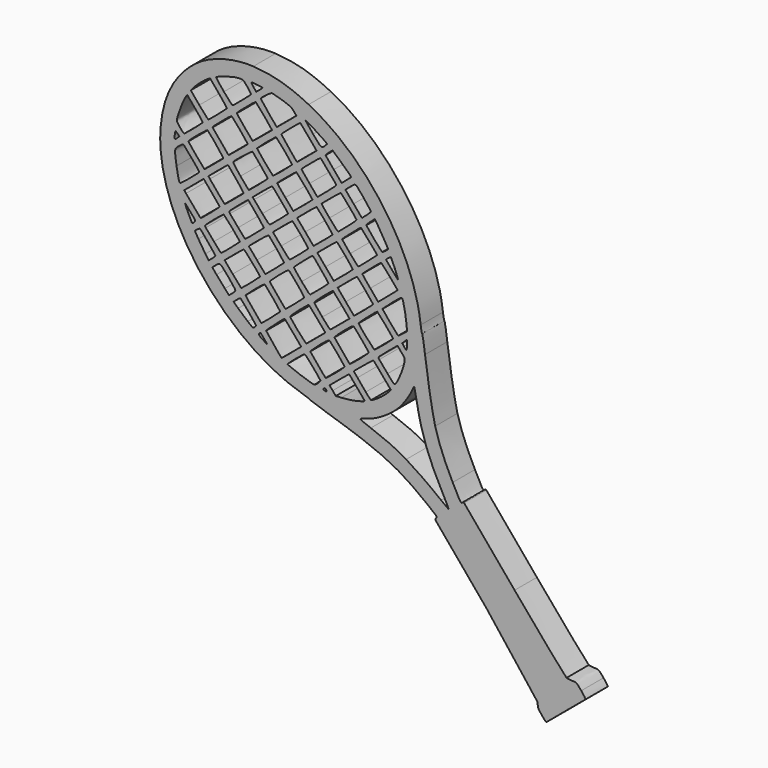
from build123d import *

# Parameters (mm, degrees)
F1_DEPTH = 3.81
F3_DEPTH = 2.286


# Not quite as in the source:
# - ends of sketch curves that miss each other by under 0.0002 mm in the source are joined


with BuildPart() as f1:
    # F0 (on Front) → F1 (new body)
    with BuildSketch(Plane.XZ):
        with BuildLine():
            add(Edge.make_bspline(
                [(8.2997352098, -34.5929658476), (7.7513746128, -33.9233854077), (7.7314698476, -33.8750955906), (7.7314698476, -33.2143245333)],
                knots=[0, 0, 0, 0, 1, 1, 1, 1], degree=3))
            add(Edge.make_bspline(
                [(9.1003873793, -35.0805100101), (8.8696736589, -35.2853643221), (8.8639067545, -35.2818536003), (8.2997352098, -34.5929658476)],
                knots=[0, 0, 0, 0, 1, 1, 1, 1], degree=3))
            add(Edge.make_bspline(
                [(11.762339667, -32.8505821788), (10.4260785287, -33.9635549553), (9.2282001786, -34.9670228107), (9.1003873793, -35.0805100101)],
                knots=[0, 0, 0, 0, 1, 1, 1, 1], degree=3))
            add(Edge.make_bspline(
                [(14.2754598273, -30.7550159293), (14.2295046015, -30.7946045899), (13.0986005293, -31.7376082979), (11.762339667, -32.8505821788)],
                knots=[0, 0, 0, 0, 1, 1, 1, 1], degree=3))
            add(Edge.make_bspline(
                [(13.6903266566, -29.8886373949), (14.0581054024, -30.3255582534), (14.3214150531, -30.715428373), (14.2754598273, -30.7550159293)],
                knots=[0, 0, 0, 0, 1, 1, 1, 1], degree=3))
            add(Edge.make_bspline(
                [(12.4820044892, -29.094235834), (13.0159091733, -29.094235834), (13.0287383819, -29.1026730513), (13.6903266566, -29.8886373949)],
                knots=[0, 0, 0, 0, 1, 1, 1, 1], degree=3))
            add(Edge.make_bspline(
                [(11.6782093458, -28.9938020258), (11.8234984493, -29.0490403994), (12.1852054908, -29.094235834), (12.4820044892, -29.094235834)],
                knots=[0, 0, 0, 0, 1, 1, 1, 1], degree=3))
            add(Edge.make_bspline(
                [(4.5755850213, -20.7461106445), (8.4195138787, -25.3257184718), (11.5297231553, -28.9373477652), (11.6782093458, -28.9938020258)],
                knots=[0, 0, 0, 0, 1, 1, 1, 1], degree=3))
            add(Edge.make_bspline(
                [(-2.3372866715, -12.4882117764), (-2.29636175, -12.5490646543), (0.8144303461, -16.2651199732), (4.5755850213, -20.7461106445)],
                knots=[0, 0, 0, 0, 1, 1, 1, 1], degree=3))
            add(Edge.make_bspline(
                [(-2.5711135485, -12.5098724545), (-2.4676648708, -12.4240182463), (-2.3855720713, -12.4164137072), (-2.3372866715, -12.4882117764)],
                knots=[0, 0, 0, 0, 1, 1, 1, 1], degree=3))
            add(Edge.make_bspline(
                [(-3.8997787065, -10.5213915001), (-2.8158337124, -12.6554707755), (-2.7911184082, -12.6924609057), (-2.5711135485, -12.5098724545)],
                knots=[0, 0, 0, 0, 1, 1, 1, 1], degree=3))
            add(Edge.make_bspline(
                [(-6.2964641631, -4.5285276805), (-5.8849079653, -6.160072376), (-5.0329179786, -8.2904553992), (-3.8997787065, -10.5213915001)],
                knots=[0, 0, 0, 0, 1, 1, 1, 1], degree=3))
            add(Edge.make_bspline(
                [(-7.6845741555, 3.6496770316), (-7.3087038532, 0.6771117347), (-6.6898074566, -2.9691863499), (-6.2964641631, -4.5285276805)],
                knots=[0, 0, 0, 0, 1, 1, 1, 1], degree=3))
            add(Edge.make_bspline(
                [(-8.0770936056, 6.0321583664), (-8.0224924406, 5.9973150884), (-7.8458586329, 4.9251987638), (-7.6845741555, 3.6496770316)],
                knots=[0, 0, 0, 0, 1, 1, 1, 1], degree=3))
            add(Edge.make_bspline(
                [(-8.2824426653, 7.0255534654), (-8.2241010743, 6.5140294943), (-8.1316947705, 6.0670016445), (-8.0770936056, 6.0321583664)],
                knots=[0, 0, 0, 0, 1, 1, 1, 1], degree=3))
            add(Edge.make_bspline(
                [(-23.6116230864, 28.5920330862), (-15.7062552337, 24.6627576065), (-9.2595784513, 15.5929903982), (-8.2824426653, 7.0255534654)],
                knots=[0, 0, 0, 0, 1, 1, 1, 1], degree=3))
            add(Edge.make_bspline(
                [(-31.18296548, 30.720503517), (-28.5010534859, 30.5700558668), (-26.4066644712, 29.9812772439), (-23.6116230864, 28.5920330862)],
                knots=[0, 0, 0, 0, 1, 1, 1, 1], degree=3))
            add(Edge.make_bspline(
                [(-39.037660333, 28.5157038779), (-37.1002587783, 29.9942754177), (-33.9583759779, 30.8761964053), (-31.18296548, 30.720503517)],
                knots=[0, 0, 0, 0, 1, 1, 1, 1], degree=3))
            add(Edge.make_bspline(
                [(-43.8690793415, 19.252351537), (-43.5308540477, 23.2937424781), (-41.9774231865, 26.2721580575), (-39.037660333, 28.5157038779)],
                knots=[0, 0, 0, 0, 1, 1, 1, 1], degree=3))
            add(Edge.make_bspline(
                [(-37.0432589699, 1.8827205194), (-41.7803909702, 7.222862873), (-44.332349939, 13.7168227214), (-43.8690793415, 19.252351537)],
                knots=[0, 0, 0, 0, 1, 1, 1, 1], degree=3))
            add(Edge.make_bspline(
                [(-24.2946169348, -6.5716153216), (-28.8978644315, -5.240519494), (-33.3340793205, -2.2986186231), (-37.0432589699, 1.8827205194)],
                knots=[0, 0, 0, 0, 1, 1, 1, 1], degree=3))
            add(Edge.make_bspline(
                [(-23.4029642962, -6.9118792415), (-23.4378296612, -6.8564608592), (-23.839073459, -6.7033419296), (-24.2946169348, -6.5716153216)],
                knots=[0, 0, 0, 0, 1, 1, 1, 1], degree=3))
            add(Edge.make_bspline(
                [(-21.083833874, -7.7199537327), (-22.3244913455, -7.3309306479), (-23.3681000355, -6.9672976238), (-23.4029642962, -6.9118792415)],
                knots=[0, 0, 0, 0, 1, 1, 1, 1], degree=3))
            add(Edge.make_bspline(
                [(-9.4411387547, -12.7401742533), (-12.3144916521, -10.7509732641), (-14.7058077695, -9.7198602697), (-21.083833874, -7.7199537327)],
                knots=[0, 0, 0, 0, 1, 1, 1, 1], degree=3))
            add(Edge.make_bspline(
                [(-6.1246397901, -15.2954793959), (-6.2230901896, -15.1361827446), (-8.3739665953, -13.4789696927), (-9.4411387547, -12.7401742533)],
                knots=[0, 0, 0, 0, 1, 1, 1, 1], degree=3))
            add(Edge.make_bspline(
                [(-6.1833126854, -15.5659750379), (-6.1121153815, -15.4801881949), (-6.0857126338, -15.3584647695), (-6.1246397901, -15.2954793959)],
                knots=[0, 0, 0, 0, 1, 1, 1, 1], degree=3))
            add(Edge.make_bspline(
                [(-6.2269653461, -15.8607740624), (-6.2741541284, -15.7844216628), (-6.2545099894, -15.6517618809), (-6.1833126854, -15.5659750379)],
                knots=[0, 0, 0, 0, 1, 1, 1, 1], degree=3))
            add(Edge.make_bspline(
                [(0.7951506419, -24.2645815733), (-3.0198255287, -19.7188396762), (-6.1797776681, -15.9371253576), (-6.2269653461, -15.8607740624)],
                knots=[0, 0, 0, 0, 1, 1, 1, 1], degree=3))
            Line((0.7951506419, -24.2645815733), (7.7314698476, -33.2143245333))
        make_face()
        with BuildLine():
            add(Edge.make_bspline(
                [(-22.3251561629, -4.5677750977), (-22.1226695727, -4.383651603), (-21.9813759996, -4.1739017172), (-22.0111690951, -4.1016641176)],
                knots=[0, 0, 0, 0, 1, 1, 1, 1], degree=3))
            add(Edge.make_bspline(
                [(-22.8589647687, -4.8979132524), (-22.7678560736, -4.9004642959), (-22.5276416488, -4.751897488), (-22.3251561629, -4.5677750977)],
                knots=[0, 0, 0, 0, 1, 1, 1, 1], degree=3))
            add(Edge.make_bspline(
                [(-26.4969890794, -3.5927695986), (-26.5119386358, -3.7445136152), (-23.3338972792, -4.8846378873), (-22.8589647687, -4.8979132524)],
                knots=[0, 0, 0, 0, 1, 1, 1, 1], degree=3))
            add(Edge.make_bspline(
                [(-24.2965440218, -1.7282715653), (-24.7322280107, -2.0422398592), (-26.4910565229, -3.5325439903), (-26.4969890794, -3.5927695986)],
                knots=[0, 0, 0, 0, 1, 1, 1, 1], degree=3))
            add(Edge.make_bspline(
                [(-23.0811739066, -2.7774019944), (-23.9946904234, -1.7046363132), (-24.1171073793, -1.598963479), (-24.2965440218, -1.7282715653)],
                knots=[0, 0, 0, 0, 1, 1, 1, 1], degree=3))
            add(Edge.make_bspline(
                [(-22.0111690951, -4.1016641176), (-22.0409621905, -4.029426518), (-22.5224644662, -3.4335082865), (-23.0811739066, -2.7774019944)],
                knots=[0, 0, 0, 0, 1, 1, 1, 1], degree=3))
        make_face(mode=Mode.SUBTRACT)
        with BuildLine():
            add(Edge.make_bspline(
                [(-21.2062596646, -5.0123225822), (-21.3076918032, -4.8227944093), (-21.356739203, -4.8079409312), (-21.4969383674, -4.9242961218)],
                knots=[0, 0, 0, 0, 1, 1, 1, 1], degree=3))
            add(Edge.make_bspline(
                [(-21.4616279502, -5.1445339989), (-21.1260067086, -5.2766073721), (-21.0780945784, -5.2518015114), (-21.2062596646, -5.0123225822)],
                knots=[0, 0, 0, 0, 1, 1, 1, 1], degree=3))
            add(Edge.make_bspline(
                [(-21.4969383674, -4.9242961218), (-21.6464195753, -5.0483541386), (-21.642405271, -5.0733952254), (-21.4616279502, -5.1445339989)],
                knots=[0, 0, 0, 0, 1, 1, 1, 1], degree=3))
        make_face(mode=Mode.SUBTRACT)
        with BuildLine():
            add(Edge.make_bspline(
                [(-17.7237474053, -5.1188148425), (-17.3593126247, -5.0553325124), (-16.7976921234, -4.9281966783), (-16.4757018469, -4.8362906441)],
                knots=[0, 0, 0, 0, 1, 1, 1, 1], degree=3))
            add(Edge.make_bspline(
                [(-19.1398128585, -5.2706328504), (-18.7254118607, -5.2506154418), (-18.0881821859, -5.1822971726), (-17.7237474053, -5.1188148425)],
                knots=[0, 0, 0, 0, 1, 1, 1, 1], degree=3))
            Line((-19.1398128585, -5.2706328504), (-19.8932696196, -5.3070299458))
            Line((-19.8932696196, -5.3070299458), (-20.318166339, -4.7995379486))
            Line((-20.318166339, -4.7995379486), (-20.7430630585, -4.292044847))
            Line((-20.7430630585, -4.292044847), (-19.42421997, -3.1924887921))
            add(Edge.make_bspline(
                [(-18.0720807947, -2.0929316329), (-18.0903941946, -2.0929316329), (-18.6988556087, -2.587732465), (-19.42421997, -3.1924887921)],
                knots=[0, 0, 0, 0, 1, 1, 1, 1], degree=3))
            add(Edge.make_bspline(
                [(-16.0339627188, -4.4872891242), (-16.4122173081, -4.0084759355), (-18.0427625688, -2.0929316329), (-18.0720807947, -2.0929316329)],
                knots=[0, 0, 0, 0, 1, 1, 1, 1], degree=3))
            add(Edge.make_bspline(
                [(-16.4757018469, -4.8362906441), (-15.9562795801, -4.6880319492), (-15.9064679717, -4.6486774103), (-16.0339627188, -4.4872891242)],
                knots=[0, 0, 0, 0, 1, 1, 1, 1], degree=3))
        make_face(mode=Mode.SUBTRACT)
        with BuildLine():
            add(Edge.make_bspline(
                [(-5.167468404, -12.4575374113), (-7.2681566187, -8.5610946064), (-8.1812104137, -6.0118644811), (-8.8500796535, -2.1757577194)],
                knots=[0, 0, 0, 0, 1, 1, 1, 1], degree=3))
            add(Edge.make_bspline(
                [(-4.4481437209, -13.9228357947), (-4.4228939124, -13.8975848818), (-4.7465904063, -13.2382008854), (-5.167468404, -12.4575374113)],
                knots=[0, 0, 0, 0, 1, 1, 1, 1], degree=3))
            add(Edge.make_bspline(
                [(-5.4767266545, -13.1803639813), (-4.9362566226, -13.613974005), (-4.4733946338, -13.9480856032), (-4.4481437209, -13.9228357947)],
                knots=[0, 0, 0, 0, 1, 1, 1, 1], degree=3))
            add(Edge.make_bspline(
                [(-10.2637354198, -9.8169479039), (-8.8669960534, -10.6556647342), (-6.9079779945, -12.0320973528), (-5.4767266545, -13.1803639813)],
                knots=[0, 0, 0, 0, 1, 1, 1, 1], degree=3))
            add(Edge.make_bspline(
                [(-15.1009213326, -7.6057630638), (-12.9494187617, -8.3928052508), (-11.6341140036, -8.9940607954), (-10.2637354198, -9.8169479039)],
                knots=[0, 0, 0, 0, 1, 1, 1, 1], degree=3))
            add(Edge.make_bspline(
                [(-16.5641821942, -7.0017709453), (-16.5641821942, -7.0395639364), (-15.9057148065, -7.3113605002), (-15.1009213326, -7.6057630638)],
                knots=[0, 0, 0, 0, 1, 1, 1, 1], degree=3))
            add(Edge.make_bspline(
                [(-15.8739648067, -6.7437952946), (-16.2535843698, -6.8478889114), (-16.5641821942, -6.9639779542), (-16.5641821942, -7.0017709453)],
                knots=[0, 0, 0, 0, 1, 1, 1, 1], degree=3))
            add(Edge.make_bspline(
                [(-10.8493257905, -3.4452983038), (-11.9459498019, -4.8390581397), (-14.1111131554, -6.2604112102), (-15.8739648067, -6.7437952946)],
                knots=[0, 0, 0, 0, 1, 1, 1, 1], degree=3))
            add(Edge.make_bspline(
                [(-9.3778618333, -1.0714098993), (-9.550148928, -1.5701631922), (-10.2043159853, -2.6255199343), (-10.8493257905, -3.4452983038)],
                knots=[0, 0, 0, 0, 1, 1, 1, 1], degree=3))
            add(Edge.make_bspline(
                [(-9.1795474691, -0.7124968578), (-9.2204304254, -0.7124968578), (-9.3096716684, -0.8740077265), (-9.3778618333, -1.0714098993)],
                knots=[0, 0, 0, 0, 1, 1, 1, 1], degree=3))
            add(Edge.make_bspline(
                [(-8.8500796535, -2.1757577194), (-8.9904047136, -1.3709642455), (-9.1386656172, -0.7124968578), (-9.1795474691, -0.7124968578)],
                knots=[0, 0, 0, 0, 1, 1, 1, 1], degree=3))
        make_face(mode=Mode.SUBTRACT)
        with BuildLine():
            add(Edge.make_bspline(
                [(-29.7059212532, -1.5959751138), (-29.9601896084, -1.2922794633), (-30.1823623028, -1.0438012038), (-30.1996387201, -1.0438012038)],
                knots=[0, 0, 0, 0, 1, 1, 1, 1], degree=3))
            add(Edge.make_bspline(
                [(-29.2829814381, -2.1481490239), (-29.2613295948, -2.1481490239), (-29.4516528981, -1.8996707644), (-29.7059212532, -1.5959751138)],
                knots=[0, 0, 0, 0, 1, 1, 1, 1], degree=3))
            add(Edge.make_bspline(
                [(-29.9077684261, -1.7539034782), (-29.5857869843, -1.9707388596), (-29.3046332815, -2.1481490239), (-29.2829814381, -2.1481490239)],
                knots=[0, 0, 0, 0, 1, 1, 1, 1], degree=3))
            add(Edge.make_bspline(
                [(-30.3621203105, -1.2017295682), (-30.469489423, -1.3311017066), (-30.38733478, -1.4309446887), (-29.9077684261, -1.7539034782)],
                knots=[0, 0, 0, 0, 1, 1, 1, 1], degree=3))
            add(Edge.make_bspline(
                [(-30.1996387201, -1.0438012038), (-30.2169151374, -1.0438012038), (-30.2900317979, -1.1148692991), (-30.3621203105, -1.2017295682)],
                knots=[0, 0, 0, 0, 1, 1, 1, 1], degree=3))
        make_face(mode=Mode.SUBTRACT)
        with BuildLine():
            add(Edge.make_bspline(
                [(-30.8102690733, -0.3623733205), (-30.8102690733, -0.284547721), (-32.367984804, 1.627009886), (-32.8436914623, 2.1329491702)],
                knots=[0, 0, 0, 0, 1, 1, 1, 1], degree=3))
            add(Edge.make_bspline(
                [(-31.0166694722, -0.6441807973), (-30.9031491424, -0.5414466326), (-30.8102690733, -0.4146332681), (-30.8102690733, -0.3623733205)],
                knots=[0, 0, 0, 0, 1, 1, 1, 1], degree=3))
            add(Edge.make_bspline(
                [(-31.9277564238, -0.2530219037), (-31.2574349665, -0.8027850225), (-31.2130037407, -0.8218604224), (-31.0166694722, -0.6441807973)],
                knots=[0, 0, 0, 0, 1, 1, 1, 1], degree=3))
            add(Edge.make_bspline(
                [(-33.2583674426, 0.9097282465), (-32.9141090967, 0.5880869439), (-32.3153339173, 0.0648502597), (-31.9277564238, -0.2530219037)],
                knots=[0, 0, 0, 0, 1, 1, 1, 1], degree=3))
            Line((-33.2583674426, 0.9097282465), (-33.8842908044, 1.4945290085))
            Line((-33.8842908044, 1.4945290085), (-33.4297092156, 1.8836338151))
            add(Edge.make_bspline(
                [(-32.8436914623, 2.1329491702), (-32.9484598356, 2.2443756566), (-33.0673627567, 2.1937899003), (-33.4297092156, 1.8836338151)],
                knots=[0, 0, 0, 0, 1, 1, 1, 1], degree=3))
        make_face(mode=Mode.SUBTRACT)
        with BuildLine():
            add(Edge.make_bspline(
                [(-33.6396777623, 2.9654474179), (-33.6470106318, 3.0551458609), (-34.1163595597, 3.6766750227), (-34.6826856871, 4.3466254191)],
                knots=[0, 0, 0, 0, 1, 1, 1, 1], degree=3))
            add(Edge.make_bspline(
                [(-34.0680951426, 2.4399390903), (-33.8251386222, 2.6392705588), (-33.6323515189, 2.8757500792), (-33.6396777623, 2.9654474179)],
                knots=[0, 0, 0, 0, 1, 1, 1, 1], degree=3))
            Line((-34.0680951426, 2.4399390903), (-34.5098342706, 2.0775164314))
            Line((-34.5098342706, 2.0775164314), (-35.0750350675, 2.6979467672))
            add(Edge.make_bspline(
                [(-36.2161024526, 4.0080588818), (-35.8993754978, 3.6287341795), (-35.3858957267, 3.0391836175), (-35.0750350675, 2.6979467672)],
                knots=[0, 0, 0, 0, 1, 1, 1, 1], degree=3))
            Line((-36.2161024526, 4.0080588818), (-36.7919668321, 4.6977395563))
            Line((-36.7919668321, 4.6977395563), (-36.4331973558, 5.0019719199))
            add(Edge.make_bspline(
                [(-34.6826856871, 4.3466254191), (-35.8100944983, 5.6803186727), (-35.6874080816, 5.6343888469), (-36.4331973558, 5.0019719199)],
                knots=[0, 0, 0, 0, 1, 1, 1, 1], degree=3))
        make_face(mode=Mode.SUBTRACT)
        with BuildLine():
            add(Edge.make_bspline(
                [(-28.7601798671, 1.2379128099), (-28.0655550274, 1.824723485), (-27.4972256131, 2.3472920386), (-27.4972256131, 2.3991776123)],
                knots=[0, 0, 0, 0, 1, 1, 1, 1], degree=3))
            add(Edge.make_bspline(
                [(-30.0675995817, 0.1709858157), (-30.0431437992, 0.1709858157), (-29.4548047068, 0.6511032392), (-28.7601798671, 1.2379128099)],
                knots=[0, 0, 0, 0, 1, 1, 1, 1], degree=3))
            add(Edge.make_bspline(
                [(-32.2265962569, 2.8187060969), (-32.2588509437, 2.7268596974), (-30.1747478246, 0.1709858157), (-30.0675995817, 0.1709858157)],
                knots=[0, 0, 0, 0, 1, 1, 1, 1], degree=3))
            add(Edge.make_bspline(
                [(-30.9315783683, 3.9824424298), (-31.6240972167, 3.3985991373), (-32.2068549353, 2.874917401), (-32.2265962569, 2.8187060969)],
                knots=[0, 0, 0, 0, 1, 1, 1, 1], degree=3))
            add(Edge.make_bspline(
                [(-29.5358318107, 4.8990036335), (-29.6469899405, 5.0169579198), (-29.9071212782, 4.8461351903), (-30.9315783683, 3.9824424298)],
                knots=[0, 0, 0, 0, 1, 1, 1, 1], degree=3))
            add(Edge.make_bspline(
                [(-27.4972256131, 2.3991776123), (-27.4972256131, 2.4771224814), (-29.0637286393, 4.3980339145), (-29.5358318107, 4.8990036335)],
                knots=[0, 0, 0, 0, 1, 1, 1, 1], degree=3))
        make_face(mode=Mode.SUBTRACT)
        with BuildLine():
            add(Edge.make_bspline(
                [(-31.5230924608, 4.5539832875), (-30.827343395, 5.1424582148), (-30.2580951633, 5.6579445859), (-30.2580951633, 5.6995100291)],
                knots=[0, 0, 0, 0, 1, 1, 1, 1], degree=3))
            add(Edge.make_bspline(
                [(-32.8367550536, 3.4840292759), (-32.8099889755, 3.4840292759), (-32.2188404222, 3.9655083603), (-31.5230924608, 4.5539832875)],
                knots=[0, 0, 0, 0, 1, 1, 1, 1], degree=3))
            add(Edge.make_bspline(
                [(-33.9951341951, 4.7936576862), (-33.3847909724, 4.0733622814), (-32.8635200274, 3.4840292759), (-32.8367550536, 3.4840292759)],
                knots=[0, 0, 0, 0, 1, 1, 1, 1], degree=3))
            Line((-33.9951341951, 4.7936576862), (-35.1048491456, 6.1032849921))
            Line((-35.1048491456, 6.1032849921), (-33.849294022, 7.1652523603))
            add(Edge.make_bspline(
                [(-32.4846790294, 8.257581563), (-32.5446627856, 8.2408827197), (-33.1587398084, 7.7493352962), (-33.849294022, 7.1652523603)],
                knots=[0, 0, 0, 0, 1, 1, 1, 1], degree=3))
            add(Edge.make_bspline(
                [(-30.2580951633, 5.6995100291), (-30.2580951633, 5.8507449413), (-32.3787168561, 8.2870797977), (-32.4846790294, 8.257581563)],
                knots=[0, 0, 0, 0, 1, 1, 1, 1], degree=3))
        make_face(mode=Mode.SUBTRACT)
        with BuildLine():
            add(Edge.make_bspline(
                [(-36.3650513649, 6.2009877481), (-36.331113652, 6.3028008867), (-38.3581286149, 8.7813626906), (-38.4917359272, 8.8014220644)],
                knots=[0, 0, 0, 0, 1, 1, 1, 1], degree=3))
            add(Edge.make_bspline(
                [(-36.8425813014, 5.7318861942), (-36.5988683027, 5.9331049931), (-36.3839798865, 6.1442010789), (-36.3650513649, 6.2009877481)],
                knots=[0, 0, 0, 0, 1, 1, 1, 1], degree=3))
            Line((-36.8425813014, 5.7318861942), (-37.2856942381, 5.3660345353))
            Line((-37.2856942381, 5.3660345353), (-37.7394453574, 6.0094518709))
            add(Edge.make_bspline(
                [(-38.6931402566, 7.498489315), (-38.4181709015, 7.0333987523), (-37.9890080865, 6.3633312951), (-37.7394453574, 6.0094518709)],
                knots=[0, 0, 0, 0, 1, 1, 1, 1], degree=3))
            Line((-38.6931402566, 7.498489315), (-39.1930840365, 8.3441094234))
            Line((-39.1930840365, 8.3441094234), (-38.8768220121, 8.577931883))
            add(Edge.make_bspline(
                [(-38.4917359272, 8.8014220644), (-38.5295885531, 8.8071094557), (-38.7028772913, 8.7065353954), (-38.8768220121, 8.577931883)],
                knots=[0, 0, 0, 0, 1, 1, 1, 1], degree=3))
        make_face(mode=Mode.SUBTRACT)
        with BuildLine():
            add(Edge.make_bspline(
                [(-39.2633989665, 9.3316923398), (-39.0768348632, 9.5378442604), (-39.0772887501, 9.5583972777), (-39.2738902708, 9.8059743894)],
                knots=[0, 0, 0, 0, 1, 1, 1, 1], degree=3))
            add(Edge.make_bspline(
                [(-39.5360017042, 9.1162031584), (-39.4933286, 9.1162031584), (-39.3706565398, 9.2131737318), (-39.2633989665, 9.3316923398)],
                knots=[0, 0, 0, 0, 1, 1, 1, 1], degree=3))
            add(Edge.make_bspline(
                [(-40.4954104989, 11.1739598515), (-40.5572429334, 11.1121263127), (-39.6266653471, 9.1162031584), (-39.5360017042, 9.1162031584)],
                knots=[0, 0, 0, 0, 1, 1, 1, 1], degree=3))
            add(Edge.make_bspline(
                [(-39.2738902708, 9.8059743894), (-39.8387951025, 10.5173466638), (-40.4582701774, 11.2110990687), (-40.4954104989, 11.1739598515)],
                knots=[0, 0, 0, 0, 1, 1, 1, 1], degree=3))
        make_face(mode=Mode.SUBTRACT)
        with BuildLine():
            add(Edge.make_bspline(
                [(-37.0448315612, 11.180070208), (-36.3490824954, 11.7685451353), (-35.7808182376, 12.2779255673), (-35.782019768, 12.3120267236)],
                knots=[0, 0, 0, 0, 1, 1, 1, 1], degree=3))
            add(Edge.make_bspline(
                [(-38.3976576408, 10.1169532138), (-38.3493512584, 10.1131873877), (-37.7405795226, 10.5915952808), (-37.0448315612, 11.180070208)],
                knots=[0, 0, 0, 0, 1, 1, 1, 1], degree=3))
            add(Edge.make_bspline(
                [(-40.3878481256, 12.4242958274), (-39.5602443475, 11.3838731808), (-38.4724904578, 10.1227775442), (-38.3976576408, 10.1169532138)],
                knots=[0, 0, 0, 0, 1, 1, 1, 1], degree=3))
            Line((-40.3878481256, 12.4242958274), (-40.6336880982, 12.7333541909))
            Line((-40.6336880982, 12.7333541909), (-39.3042311228, 13.8503140772))
            Line((-39.3042311228, 13.8503140772), (-37.9747741474, 14.9672746538))
            Line((-37.9747741474, 14.9672746538), (-36.8794897099, 13.6706521478))
            add(Edge.make_bspline(
                [(-35.782019768, 12.3120267236), (-35.7832235072, 12.34612788), (-36.2770834349, 12.9575091897), (-36.8794897099, 13.6706521478)],
                knots=[0, 0, 0, 0, 1, 1, 1, 1], degree=3))
        make_face(mode=Mode.SUBTRACT)
        with BuildLine():
            add(Edge.make_bspline(
                [(-34.283962011, 7.8670267478), (-33.5882129452, 8.455501675), (-33.0198581309, 8.964882107), (-33.0209503309, 8.9989832634)],
                knots=[0, 0, 0, 0, 1, 1, 1, 1], degree=3))
            add(Edge.make_bspline(
                [(-35.5996554995, 6.7970727362), (-35.5717718214, 6.7970727362), (-34.9797099724, 7.2785518205), (-34.283962011, 7.8670267478)],
                knots=[0, 0, 0, 0, 1, 1, 1, 1], degree=3))
            add(Edge.make_bspline(
                [(-36.5638582681, 7.8738118608), (-36.06143081, 7.2816053423), (-35.6275391776, 6.7970727362), (-35.5996554995, 6.7970727362)],
                knots=[0, 0, 0, 0, 1, 1, 1, 1], degree=3))
            add(Edge.make_bspline(
                [(-37.6775543925, 9.1783525406), (-37.5674487062, 9.0530620718), (-37.0662857263, 8.4660183793), (-36.5638582681, 7.8738118608)],
                knots=[0, 0, 0, 0, 1, 1, 1, 1], degree=3))
            add(Edge.make_bspline(
                [(-36.6161778505, 10.4732091945), (-37.8614503915, 9.4199396698), (-37.8751608697, 9.4032121133), (-37.6775543925, 9.1783525406)],
                knots=[0, 0, 0, 0, 1, 1, 1, 1], degree=3))
            add(Edge.make_bspline(
                [(-35.2518279014, 11.5706250233), (-35.3083572576, 11.5539261799), (-35.9223150108, 11.0600894435), (-36.6161778505, 10.4732091945)],
                knots=[0, 0, 0, 0, 1, 1, 1, 1], degree=3))
            add(Edge.make_bspline(
                [(-33.0209503309, 8.9989832634), (-33.0254892004, 9.1407252017), (-35.1575618758, 11.5984700492), (-35.2518279014, 11.5706250233)],
                knots=[0, 0, 0, 0, 1, 1, 1, 1], degree=3))
        make_face(mode=Mode.SUBTRACT)
        with BuildLine():
            add(Edge.make_bspline(
                [(-31.0120510896, 10.6125458633), (-30.3240490238, 11.1925780514), (-29.7484055139, 11.7028861356), (-29.7328430444, 11.7465630919)],
                knots=[0, 0, 0, 0, 1, 1, 1, 1], degree=3))
            add(Edge.make_bspline(
                [(-32.300136987, 9.5579422864), (-32.2796910914, 9.5579422864), (-31.7000520511, 10.0325136751), (-31.0120510896, 10.6125458633)],
                knots=[0, 0, 0, 0, 1, 1, 1, 1], degree=3))
            add(Edge.make_bspline(
                [(-33.2508148079, 10.634681411), (-32.7483873497, 10.0424748925), (-32.3205817782, 9.5579422864), (-32.300136987, 9.5579422864)],
                knots=[0, 0, 0, 0, 1, 1, 1, 1], degree=3))
            add(Edge.make_bspline(
                [(-34.3680161322, 11.9429536821), (-34.2559833589, 11.8156102307), (-33.753242266, 11.2268879295), (-33.2508148079, 10.634681411)],
                knots=[0, 0, 0, 0, 1, 1, 1, 1], degree=3))
            add(Edge.make_bspline(
                [(-33.2359381384, 13.3069579704), (-34.5623548442, 12.1824226721), (-34.5702873746, 12.1728645418), (-34.3680161322, 11.9429536821)],
                knots=[0, 0, 0, 0, 1, 1, 1, 1], degree=3))
            add(Edge.make_bspline(
                [(-31.8655518241, 14.400642622), (-31.8845874675, 14.4219764132), (-32.5012619163, 13.9298182855), (-33.2359381384, 13.3069579704)],
                knots=[0, 0, 0, 0, 1, 1, 1, 1], degree=3))
            add(Edge.make_bspline(
                [(-29.7328430444, 11.7465630919), (-29.7122911315, 11.8042442829), (-31.1930481756, 13.6469937044), (-31.8655518241, 14.400642622)],
                knots=[0, 0, 0, 0, 1, 1, 1, 1], degree=3))
        make_face(mode=Mode.SUBTRACT)
        with BuildLine():
            add(Edge.make_bspline(
                [(-25.7471512661, 0.4010656405), (-26.3607898627, 1.1248673496), (-26.8750349469, 1.7170683464), (-26.8899160338, 1.7170683464)],
                knots=[0, 0, 0, 0, 1, 1, 1, 1], degree=3))
            Line((-25.7471512661, 0.4010656405), (-24.6314441243, -0.914935961))
            Line((-24.6314441243, -0.914935961), (-25.9456136128, -2.0284995637))
            add(Edge.make_bspline(
                [(-27.2956788229, -3.141608175), (-27.2759363969, -3.1418290446), (-26.6684070524, -2.6409587169), (-25.9456136128, -2.0284995637)],
                knots=[0, 0, 0, 0, 1, 1, 1, 1], degree=3))
            add(Edge.make_bspline(
                [(-29.4165114461, -0.5442682413), (-29.404810881, -0.6707812232), (-27.3882364224, -3.140436462), (-27.2956788229, -3.141608175)],
                knots=[0, 0, 0, 0, 1, 1, 1, 1], degree=3))
            add(Edge.make_bspline(
                [(-26.8899160338, 1.7170683464), (-27.0223317548, 1.7170683464), (-29.4266350026, -0.4348163288), (-29.4165114461, -0.5442682413)],
                knots=[0, 0, 0, 0, 1, 1, 1, 1], degree=3))
        make_face(mode=Mode.SUBTRACT)
        with BuildLine():
            add(Edge.make_bspline(
                [(-25.4903119892, 3.9864589428), (-24.8023099234, 4.5664911309), (-24.22279457, 5.0884158498), (-24.2024988658, 5.1462925104)],
                knots=[0, 0, 0, 0, 1, 1, 1, 1], degree=3))
            add(Edge.make_bspline(
                [(-26.7701230083, 2.9318553659), (-26.7542292345, 2.9318553659), (-26.1783129507, 3.4064267546), (-25.4903119892, 3.9864589428)],
                knots=[0, 0, 0, 0, 1, 1, 1, 1], degree=3))
            add(Edge.make_bspline(
                [(-28.9328777792, 5.5574467255), (-28.9328777792, 5.4692192738), (-26.8427979297, 2.9318553659), (-26.7701230083, 2.9318553659)],
                knots=[0, 0, 0, 0, 1, 1, 1, 1], degree=3))
            add(Edge.make_bspline(
                [(-27.6528017166, 6.7385235278), (-28.3568433301, 6.1437571311), (-28.9328777792, 5.6122731774), (-28.9328777792, 5.5574467255)],
                knots=[0, 0, 0, 0, 1, 1, 1, 1], degree=3))
            add(Edge.make_bspline(
                [(-26.1811522289, 7.6121896535), (-26.3666594714, 7.8133377742), (-26.413258532, 7.7856727569), (-27.6528017166, 6.7385235278)],
                knots=[0, 0, 0, 0, 1, 1, 1, 1], degree=3))
            add(Edge.make_bspline(
                [(-24.2024988658, 5.1462925104), (-24.1722364224, 5.2325906664), (-25.4153267722, 6.7817918754), (-26.1811522289, 7.6121896535)],
                knots=[0, 0, 0, 0, 1, 1, 1, 1], degree=3))
        make_face(mode=Mode.SUBTRACT)
        with BuildLine():
            add(Edge.make_bspline(
                [(-22.437194458, 3.1655817472), (-23.049135672, 3.8873801694), (-23.5705601214, 4.477942314), (-23.595914843, 4.477942314)],
                knots=[0, 0, 0, 0, 1, 1, 1, 1], degree=3))
            Line((-22.437194458, 3.1655817472), (-21.3245750727, 1.8532200761))
            Line((-21.3245750727, 1.8532200761), (-22.5611177442, 0.8120420557))
            add(Edge.make_bspline(
                [(-23.913093476, -0.2977049209), (-23.8496056242, -0.2599925472), (-23.2412159927, 0.2393935371), (-22.5611177442, 0.8120420557)],
                knots=[0, 0, 0, 0, 1, 1, 1, 1], degree=3))
            add(Edge.make_bspline(
                [(-26.1226482988, 2.1894719004), (-25.998634456, 1.8662966586), (-24.0198463624, -0.3611187814), (-23.913093476, -0.2977049209)],
                knots=[0, 0, 0, 0, 1, 1, 1, 1], degree=3))
            add(Edge.make_bspline(
                [(-24.909898801, 3.4055465894), (-25.6608045187, 2.7704184885), (-26.1553016551, 2.274565213), (-26.1226482988, 2.1894719004)],
                knots=[0, 0, 0, 0, 1, 1, 1, 1], degree=3))
            add(Edge.make_bspline(
                [(-23.595914843, 4.477942314), (-23.6212695646, 4.477942314), (-24.2125627874, 3.9953644036), (-24.909898801, 3.4055465894)],
                knots=[0, 0, 0, 0, 1, 1, 1, 1], degree=3))
        make_face(mode=Mode.SUBTRACT)
        with BuildLine():
            add(Edge.make_bspline(
                [(-19.9129778108, -2.5254373088), (-19.2184457363, -1.9433377815), (-18.6653728872, -1.4239166191), (-18.6839270349, -1.3711685498)],
                knots=[0, 0, 0, 0, 1, 1, 1, 1], degree=3))
            add(Edge.make_bspline(
                [(-21.2719286034, -3.5772612422), (-21.2190369689, -3.5808614161), (-20.6075087809, -3.1075379404), (-19.9129778108, -2.5254373088)],
                knots=[0, 0, 0, 0, 1, 1, 1, 1], degree=3))
            add(Edge.make_bspline(
                [(-23.3796371572, -1.0830883775), (-23.3181735749, -1.2674802287), (-21.3720388377, -3.5704529379), (-21.2719286034, -3.5772612422)],
                knots=[0, 0, 0, 0, 1, 1, 1, 1], degree=3))
            add(Edge.make_bspline(
                [(-22.1373585031, 0.1023693726), (-22.8398783253, -0.4918327024), (-23.3989036093, -1.0252890213), (-23.3796371572, -1.0830883775)],
                knots=[0, 0, 0, 0, 1, 1, 1, 1], degree=3))
            add(Edge.make_bspline(
                [(-20.717340589, 1.0642982891), (-20.8256903624, 1.1542198103), (-21.167588717, 0.9226159855), (-22.1373585031, 0.1023693726)],
                knots=[0, 0, 0, 0, 1, 1, 1, 1], degree=3))
            add(Edge.make_bspline(
                [(-18.6839270349, -1.3711685498), (-18.7266995303, -1.2495632896), (-20.5260001814, 0.9054996987), (-20.717340589, 1.0642982891)],
                knots=[0, 0, 0, 0, 1, 1, 1, 1], degree=3))
        make_face(mode=Mode.SUBTRACT)
        with BuildLine():
            add(Edge.make_bspline(
                [(-16.6102279766, 0.2409716501), (-15.9120637021, 0.8261158643), (-15.3551896877, 1.3453691658), (-15.3727278355, 1.3948671395)],
                knots=[0, 0, 0, 0, 1, 1, 1, 1], degree=3))
            add(Edge.make_bspline(
                [(-17.9673345083, -0.8163872746), (-17.9190888651, -0.8199874485), (-17.3083911467, -0.3441725641), (-16.6102279766, 0.2409716501)],
                knots=[0, 0, 0, 0, 1, 1, 1, 1], degree=3))
            add(Edge.make_bspline(
                [(-20.0694009491, 1.6862062422), (-20.0093752277, 1.506129078), (-18.0646595774, -0.8091317094), (-17.9673345083, -0.8163872746)],
                knots=[0, 0, 0, 0, 1, 1, 1, 1], degree=3))
            add(Edge.make_bspline(
                [(-18.8299726167, 2.8774209575), (-19.5324681433, 2.2846832477), (-20.0902101751, 1.7486361289), (-20.0694009491, 1.6862062422)],
                knots=[0, 0, 0, 0, 1, 1, 1, 1], degree=3))
            add(Edge.make_bspline(
                [(-17.3309242596, 3.7544133788), (-17.5483195454, 3.9511540473), (-17.5779878496, 3.9337970126), (-18.8299726167, 2.8774209575)],
                knots=[0, 0, 0, 0, 1, 1, 1, 1], degree=3))
            add(Edge.make_bspline(
                [(-15.3727278355, 1.3948671395), (-15.4202909917, 1.529100617), (-17.0744935914, 3.5223468323), (-17.3309242596, 3.7544133788)],
                knots=[0, 0, 0, 0, 1, 1, 1, 1], degree=3))
        make_face(mode=Mode.SUBTRACT)
        with BuildLine():
            add(Edge.make_bspline(
                [(-19.1232608934, 5.9307604626), (-19.7328697248, 6.6501889544), (-20.2566420176, 7.2388118642), (-20.2872004262, 7.2388118642)],
                knots=[0, 0, 0, 0, 1, 1, 1, 1], degree=3))
            Line((-19.1232608934, 5.9307604626), (-18.0148833081, 4.6227090611))
            Line((-18.0148833081, 4.6227090611), (-19.1848846061, 3.639238736))
            add(Edge.make_bspline(
                [(-20.538546677, 2.5249451594), (-20.4375330862, 2.5968978373), (-19.8283858721, 3.098330278), (-19.1848846061, 3.639238736)],
                knots=[0, 0, 0, 0, 1, 1, 1, 1], degree=3))
            add(Edge.make_bspline(
                [(-21.7371561052, 3.597312171), (-20.8635860578, 2.5617232549), (-20.6966230239, 2.4123447513), (-20.538546677, 2.5249451594)],
                knots=[0, 0, 0, 0, 1, 1, 1, 1], degree=3))
            add(Edge.make_bspline(
                [(-22.8108648994, 4.9536235723), (-22.7785472648, 4.8694071119), (-22.2953785283, 4.2590660978), (-21.7371561052, 3.597312171)],
                knots=[0, 0, 0, 0, 1, 1, 1, 1], degree=3))
            add(Edge.make_bspline(
                [(-21.6061914973, 6.1727782874), (-22.4103996668, 5.4942194998), (-22.848265847, 5.0510899979), (-22.8108648994, 4.9536235723)],
                knots=[0, 0, 0, 0, 1, 1, 1, 1], degree=3))
            add(Edge.make_bspline(
                [(-20.2872004262, 7.2388118642), (-20.3177577303, 7.2388118642), (-20.9113038228, 6.7590964234), (-21.6061914973, 6.1727782874)],
                knots=[0, 0, 0, 0, 1, 1, 1, 1], degree=3))
        make_face(mode=Mode.SUBTRACT)
        with BuildLine():
            add(Edge.make_bspline(
                [(-28.2511815394, 7.299502403), (-27.5631794736, 7.8795345912), (-26.9862493985, 8.393702371), (-26.9691143377, 8.4420971012)],
                knots=[0, 0, 0, 0, 1, 1, 1, 1], degree=3))
            add(Edge.make_bspline(
                [(-29.5372354368, 6.2448988262), (-29.5179071412, 6.2448988262), (-28.9391825009, 6.7194702149), (-28.2511815394, 7.299502403)],
                knots=[0, 0, 0, 0, 1, 1, 1, 1], degree=3))
            add(Edge.make_bspline(
                [(-30.6866671523, 7.5599274973), (-30.0738071208, 6.8366613969), (-29.556562628, 6.2448988262), (-29.5372354368, 6.2448988262)],
                knots=[0, 0, 0, 0, 1, 1, 1, 1], degree=3))
            Line((-30.6866671523, 7.5599274973), (-31.8009574158, 8.8749561684))
            Line((-31.8009574158, 8.8749561684), (-30.4691967708, 10.0034240492))
            add(Edge.make_bspline(
                [(-29.0471899264, 11.0351344958), (-29.0968502392, 11.0883784172), (-29.7363626009, 10.6243922024), (-30.4691967708, 10.0034240492)],
                knots=[0, 0, 0, 0, 1, 1, 1, 1], degree=3))
            add(Edge.make_bspline(
                [(-26.9691143377, 8.4420971012), (-26.9452990769, 8.5093596138), (-28.4950988424, 10.4432106903), (-29.0471899264, 11.0351344958)],
                knots=[0, 0, 0, 0, 1, 1, 1, 1], degree=3))
        make_face(mode=Mode.SUBTRACT)
        with BuildLine():
            add(Edge.make_bspline(
                [(-22.0307039036, 6.8956921009), (-21.4233126026, 7.4064982459), (-20.9102049967, 7.8653602869), (-20.8904636751, 7.9153839301)],
                knots=[0, 0, 0, 0, 1, 1, 1, 1], degree=3))
            add(Edge.make_bspline(
                [(-23.3111355662, 5.8305718197), (-23.2142897842, 5.9055813323), (-22.6380952047, 6.3848848515), (-22.0307039036, 6.8956921009)],
                knots=[0, 0, 0, 0, 1, 1, 1, 1], degree=3))
            add(Edge.make_bspline(
                [(-24.5535268638, 6.9564124571), (-23.6374361123, 5.8720091586), (-23.462413548, 5.7134049334), (-23.3111355662, 5.8305718197)],
                knots=[0, 0, 0, 0, 1, 1, 1, 1], degree=3))
            add(Edge.make_bspline(
                [(-25.6198343189, 8.3260754235), (-25.6198343189, 8.2669817717), (-25.1399962954, 7.6506342098), (-24.5535268638, 6.9564124571)],
                knots=[0, 0, 0, 0, 1, 1, 1, 1], degree=3))
            add(Edge.make_bspline(
                [(-23.0571178981, 10.5518553245), (-23.1721832105, 10.5518553245), (-25.6198343189, 8.4260122752), (-25.6198343189, 8.3260754235)],
                knots=[0, 0, 0, 0, 1, 1, 1, 1], degree=3))
            add(Edge.make_bspline(
                [(-20.8904636751, 7.9153839301), (-20.8559296144, 8.0028968688), (-22.9506653943, 10.5518553245), (-23.0571178981, 10.5518553245)],
                knots=[0, 0, 0, 0, 1, 1, 1, 1], degree=3))
        make_face(mode=Mode.SUBTRACT)
        with BuildLine():
            add(Edge.make_bspline(
                [(-24.7934541582, 10.2095616133), (-24.1850291876, 10.7198001236), (-23.6726383034, 11.1735523472), (-23.6548086079, 11.217900747)],
                knots=[0, 0, 0, 0, 1, 1, 1, 1], degree=3))
            add(Edge.make_bspline(
                [(-26.0775522556, 9.1415026626), (-25.9797247083, 9.2186965752), (-25.4018802331, 9.699323103), (-24.7934541582, 10.2095616133)],
                knots=[0, 0, 0, 0, 1, 1, 1, 1], degree=3))
            add(Edge.make_bspline(
                [(-27.3752813181, 10.3227528475), (-26.4031990277, 9.1755519146), (-26.2319489156, 9.0196721154), (-26.0775522556, 9.1415026626)],
                knots=[0, 0, 0, 0, 1, 1, 1, 1], degree=3))
            Line((-27.3752813181, 10.3227528475), (-28.4951408076, 11.6443545968))
            Line((-28.4951408076, 11.6443545968), (-27.2151177537, 12.7270174431))
            add(Edge.make_bspline(
                [(-25.8351026308, 13.8096818079), (-25.8900980479, 13.8096818079), (-26.5111048532, 13.322482892), (-27.2151177537, 12.7270174431)],
                knots=[0, 0, 0, 0, 1, 1, 1, 1], degree=3))
            add(Edge.make_bspline(
                [(-23.6548086079, 11.217900747), (-23.6125187124, 11.3230898768), (-25.7043235532, 13.8096818079), (-25.8351026308, 13.8096818079)],
                knots=[0, 0, 0, 0, 1, 1, 1, 1], degree=3))
        make_face(mode=Mode.SUBTRACT)
        with BuildLine():
            add(Edge.make_bspline(
                [(-21.2687193687, 13.1470727017), (-20.7525891628, 13.5722466124), (-20.3277509738, 13.9535540332), (-20.3246333999, 13.9944215286)],
                knots=[0, 0, 0, 0, 1, 1, 1, 1], degree=3))
            add(Edge.make_bspline(
                [(-22.5744582659, 12.0707002206), (-22.3724310844, 12.2375307327), (-21.7848484702, 12.721898791), (-21.2687193687, 13.1470727017)],
                knots=[0, 0, 0, 0, 1, 1, 1, 1], degree=3))
            Line((-22.5744582659, 12.0707002206), (-22.9417798117, 11.7673712135))
            Line((-22.9417798117, 11.7673712135), (-24.0664133969, 13.0939027715))
            Line((-24.0664133969, 13.0939027715), (-25.1910469821, 14.4204336393))
            Line((-25.1910469821, 14.4204336393), (-24.880875436, 14.6815986466))
            add(Edge.make_bspline(
                [(-23.5767908518, 15.7833379971), (-24.1234430227, 15.3210215562), (-24.7102813065, 14.8252389589), (-24.880875436, 14.6815986466)],
                knots=[0, 0, 0, 0, 1, 1, 1, 1], degree=3))
            add(Edge.make_bspline(
                [(-22.505524875, 16.5972324014), (-22.5480687704, 16.6119058709), (-23.0301386808, 16.2456533338), (-23.5767908518, 15.7833379971)],
                knots=[0, 0, 0, 0, 1, 1, 1, 1], degree=3))
            add(Edge.make_bspline(
                [(-20.3246333999, 13.9944215286), (-20.3179300086, 14.0822348499), (-22.3926152495, 16.5582864712), (-22.505524875, 16.5972324014)],
                knots=[0, 0, 0, 0, 1, 1, 1, 1], degree=3))
        make_face(mode=Mode.SUBTRACT)
        with BuildLine():
            add(Edge.make_bspline(
                [(-15.849190972, 6.4286623034), (-15.2768306882, 6.9046141269), (-14.8059908907, 7.337917142), (-14.8028799429, 7.3915586286)],
                knots=[0, 0, 0, 0, 1, 1, 1, 1], degree=3))
            add(Edge.make_bspline(
                [(-17.1489200084, 5.359508944), (-17.0064304266, 5.471591413), (-16.4215523602, 5.9527104799), (-15.849190972, 6.4286623034)],
                knots=[0, 0, 0, 0, 1, 1, 1, 1], degree=3))
            Line((-17.1489200084, 5.359508944), (-17.4079933809, 5.1557225364))
            Line((-17.4079933809, 5.1557225364), (-18.5246679314, 6.4869718683))
            Line((-18.5246679314, 6.4869718683), (-19.6413413775, 7.8182200959))
            Line((-19.6413413775, 7.8182200959), (-18.3512400454, 8.9080269682))
            add(Edge.make_bspline(
                [(-16.9883511484, 9.9987581797), (-17.0283848613, 9.9982060058), (-17.6416844231, 9.5074205823), (-18.3512400454, 8.9080269682)],
                knots=[0, 0, 0, 0, 1, 1, 1, 1], degree=3))
            add(Edge.make_bspline(
                [(-14.8028799429, 7.3915586286), (-14.7960771604, 7.5088613497), (-16.8843282099, 10.0000778753), (-16.9883511484, 9.9987581797)],
                knots=[0, 0, 0, 0, 1, 1, 1, 1], degree=3))
        make_face(mode=Mode.SUBTRACT)
        with BuildLine():
            add(Edge.make_bspline(
                [(-18.5078498184, 9.8340292414), (-17.9917196126, 10.2592031522), (-17.5668814236, 10.647515037), (-17.5637638497, 10.6969445411)],
                knots=[0, 0, 0, 0, 1, 1, 1, 1], degree=3))
            add(Edge.make_bspline(
                [(-19.8106920114, 8.7599814125), (-19.6102584038, 8.9255341942), (-19.02397892, 9.4088553307), (-18.5078498184, 9.8340292414)],
                knots=[0, 0, 0, 0, 1, 1, 1, 1], degree=3))
            Line((-19.8106920114, 8.7599814125), (-20.1751157485, 8.4589770576))
            Line((-20.1751157485, 8.4589770576), (-21.295705212, 9.7906272678))
            Line((-21.295705212, 9.7906272678), (-22.4162946755, 11.1222785823))
            Line((-22.4162946755, 11.1222785823), (-21.6140323668, 11.8033718481))
            add(Edge.make_bspline(
                [(-19.7456050639, 13.3127248747), (-19.805985281, 13.3127248747), (-20.4285492167, 12.8098048774), (-21.6140323668, 11.8033718481)],
                knots=[0, 0, 0, 0, 1, 1, 1, 1], degree=3))
            add(Edge.make_bspline(
                [(-17.5637638497, 10.6969445411), (-17.5575905453, 10.7947511058), (-19.6578557948, 13.3127248747), (-19.7456050639, 13.3127248747)],
                knots=[0, 0, 0, 0, 1, 1, 1, 1], degree=3))
        make_face(mode=Mode.SUBTRACT)
        with BuildLine():
            add(Edge.make_bspline(
                [(-15.3217908966, 12.531833905), (-14.7295843781, 13.0328378588), (-14.245051772, 13.4663595347), (-14.245051772, 13.4952172476)],
                knots=[0, 0, 0, 0, 1, 1, 1, 1], degree=3))
            add(Edge.make_bspline(
                [(-16.6266661939, 11.4175524763), (-16.5011912989, 11.5294041366), (-15.9139974151, 12.0308310556), (-15.3217908966, 12.531833905)],
                knots=[0, 0, 0, 0, 1, 1, 1, 1], degree=3))
            add(Edge.make_bspline(
                [(-17.9249662042, 12.486398827), (-16.865306923, 11.226673686), (-16.8525616448, 11.2161812774), (-16.6266661939, 11.4175524763)],
                knots=[0, 0, 0, 0, 1, 1, 1, 1], degree=3))
            add(Edge.make_bspline(
                [(-19.0220474156, 13.8491865381), (-19.0072436331, 13.7993716166), (-18.513557088, 13.1861169189), (-17.9249662042, 12.486398827)],
                knots=[0, 0, 0, 0, 1, 1, 1, 1], degree=3))
            add(Edge.make_bspline(
                [(-16.4515320905, 16.073594839), (-16.5850300724, 16.073594839), (-19.0493568329, 13.9410771115), (-19.0220474156, 13.8491865381)],
                knots=[0, 0, 0, 0, 1, 1, 1, 1], degree=3))
            add(Edge.make_bspline(
                [(-14.245051772, 13.4952172476), (-14.245051772, 13.5849764297), (-16.3747202822, 16.073594839), (-16.4515320905, 16.073594839)],
                knots=[0, 0, 0, 0, 1, 1, 1, 1], degree=3))
        make_face(mode=Mode.SUBTRACT)
        with BuildLine():
            add(Edge.make_bspline(
                [(-39.9470476932, 14.3741526309), (-39.3254069923, 14.8971993672), (-38.7473471693, 15.3908306949), (-38.6624725176, 15.4711101554)],
                knots=[0, 0, 0, 0, 1, 1, 1, 1], degree=3))
            add(Edge.make_bspline(
                [(-41.1842485561, 13.4231596567), (-41.1254298868, 13.4231596567), (-40.5686894985, 13.8511069989), (-39.9470476932, 14.3741526309)],
                knots=[0, 0, 0, 0, 1, 1, 1, 1], degree=3))
            add(Edge.make_bspline(
                [(-41.6840266838, 15.300551365), (-41.4993477022, 14.0554522065), (-41.3310252161, 13.4231596567), (-41.1842485561, 13.4231596567)],
                knots=[0, 0, 0, 0, 1, 1, 1, 1], degree=3))
            add(Edge.make_bspline(
                [(-41.3652500594, 17.8218798665), (-41.9866135691, 17.3078713889), (-41.9843805778, 17.3255299105), (-41.6840266838, 15.300551365)],
                knots=[0, 0, 0, 0, 1, 1, 1, 1], degree=3))
            add(Edge.make_bspline(
                [(-40.7446838889, 18.2241584382), (-40.7869528017, 18.2502817859), (-41.0662070263, 18.0692559869), (-41.3652500594, 17.8218798665)],
                knots=[0, 0, 0, 0, 1, 1, 1, 1], degree=3))
            add(Edge.make_bspline(
                [(-39.5879943995, 16.8968684694), (-40.1819060311, 17.6007551981), (-40.7024160804, 18.1980350905), (-40.7446838889, 18.2241584382)],
                knots=[0, 0, 0, 0, 1, 1, 1, 1], degree=3))
            add(Edge.make_bspline(
                [(-38.6624725176, 15.4711101554), (-38.5319419183, 15.5945762416), (-38.6746026741, 15.8143436665), (-39.5879943995, 16.8968684694)],
                knots=[0, 0, 0, 0, 1, 1, 1, 1], degree=3))
        make_face(mode=Mode.SUBTRACT)
        with BuildLine():
            add(Edge.make_bspline(
                [(-41.8941023522, 19.1572528332), (-42.0386404993, 18.4345632023), (-41.9451905867, 18.3292525942), (-41.5410743802, 18.759414844)],
                knots=[0, 0, 0, 0, 1, 1, 1, 1], degree=3))
            Line((-41.8941023522, 19.1572528332), (-41.8240237526, 19.5076491443))
            Line((-41.8240237526, 19.5076491443), (-41.5621795714, 19.2616589804))
            Line((-41.5621795714, 19.2616589804), (-41.3003353902, 19.0156699209))
            Line((-41.3003353902, 19.0156699209), (-41.5410743802, 18.759414844))
        make_face(mode=Mode.SUBTRACT)
        with BuildLine():
            add(Edge.make_bspline(
                [(-36.5932504854, 17.189975633), (-35.9332844977, 17.7432458843), (-35.3490425356, 18.2372615251), (-35.2949339098, 18.2877887509)],
                knots=[0, 0, 0, 0, 1, 1, 1, 1], degree=3))
            add(Edge.make_bspline(
                [(-37.8632504785, 16.1850445167), (-37.82471647, 16.1844923428), (-37.2532164731, 16.6367051055), (-36.5932504854, 17.189975633)],
                knots=[0, 0, 0, 0, 1, 1, 1, 1], degree=3))
            add(Edge.make_bspline(
                [(-40.0570573013, 18.8004822264), (-40.0039028321, 18.6410177142), (-37.9448452172, 16.1862272732), (-37.8632504785, 16.1850445167)],
                knots=[0, 0, 0, 0, 1, 1, 1, 1], degree=3))
            add(Edge.make_bspline(
                [(-37.4395122199, 20.9898931928), (-37.5565178714, 21.0622064402), (-40.1014167446, 18.9335594518), (-40.0570573013, 18.8004822264)],
                knots=[0, 0, 0, 0, 1, 1, 1, 1], degree=3))
            add(Edge.make_bspline(
                [(-35.2949339098, 18.2877887509), (-35.213354632, 18.3639688722), (-37.160717404, 20.8175882904), (-37.4395122199, 20.9898931928)],
                knots=[0, 0, 0, 0, 1, 1, 1, 1], degree=3))
        make_face(mode=Mode.SUBTRACT)
        with BuildLine():
            add(Edge.make_bspline(
                [(-39.2861385925, 20.6412366436), (-38.6331929438, 21.185572445), (-38.0989646859, 21.6748239293), (-38.0989646859, 21.7284622409)],
                knots=[0, 0, 0, 0, 1, 1, 1, 1], degree=3))
            add(Edge.make_bspline(
                [(-40.5895727158, 19.5812495091), (-40.5256298727, 19.6199061002), (-39.9390842411, 20.0969008422), (-39.2861385925, 20.6412366436)],
                knots=[0, 0, 0, 0, 1, 1, 1, 1], degree=3))
            add(Edge.make_bspline(
                [(-41.6328777102, 20.8231220393), (-41.6328777102, 20.5337064344), (-40.7508174367, 19.4837676227), (-40.5895727158, 19.5812495091)],
                knots=[0, 0, 0, 0, 1, 1, 1, 1], degree=3))
            add(Edge.make_bspline(
                [(-40.5951982636, 23.7366411713), (-40.9768829572, 23.0632147021), (-41.6328777102, 21.2213606306), (-41.6328777102, 20.8231220393)],
                knots=[0, 0, 0, 0, 1, 1, 1, 1], degree=3))
            Line((-40.5951982636, 23.7366411713), (-40.2341770221, 24.3736111863))
            Line((-40.2341770221, 24.3736111863), (-39.166570854, 23.0997988465))
            add(Edge.make_bspline(
                [(-38.0989646859, 21.7284622409), (-38.0989646859, 21.7821005526), (-38.5793880137, 22.3992019699), (-39.166570854, 23.0997988465)],
                knots=[0, 0, 0, 0, 1, 1, 1, 1], degree=3))
        make_face(mode=Mode.SUBTRACT)
        with BuildLine():
            add(Edge.make_bspline(
                [(-33.8269099961, 13.8767035727), (-33.1699533561, 14.4298482045), (-32.5879024202, 14.9241344105), (-32.5334635944, 14.975117732)],
                knots=[0, 0, 0, 0, 1, 1, 1, 1], degree=3))
            add(Edge.make_bspline(
                [(-35.0969099892, 12.8766400075), (-35.0553677372, 12.8735257467), (-34.4838677403, 13.3235585268), (-33.8269099961, 13.8767035727)],
                knots=[0, 0, 0, 0, 1, 1, 1, 1], degree=3))
            add(Edge.make_bspline(
                [(-37.1139040999, 15.2315053306), (-36.4371520253, 14.3711543266), (-35.1611896584, 12.8814527553), (-35.0969099892, 12.8766400075)],
                knots=[0, 0, 0, 0, 1, 1, 1, 1], degree=3))
            Line((-37.1139040999, 15.2315053306), (-37.3246324379, 15.4994024422))
            Line((-37.3246324379, 15.4994024422), (-35.9938966278, 16.6270034099))
            add(Edge.make_bspline(
                [(-34.6330518786, 17.7147503975), (-34.6496126785, 17.736669493), (-35.2619923187, 17.2471830588), (-35.9938966278, 16.6270034099)],
                knots=[0, 0, 0, 0, 1, 1, 1, 1], degree=3))
            add(Edge.make_bspline(
                [(-33.5187130238, 16.3713568287), (-34.1150398641, 17.0883049553), (-34.6164921831, 17.6928324063), (-34.6330518786, 17.7147503975)],
                knots=[0, 0, 0, 0, 1, 1, 1, 1], degree=3))
            add(Edge.make_bspline(
                [(-32.5334635944, 14.975117732), (-32.477098786, 15.0279044534), (-32.9012953489, 15.6290517719), (-33.5187130238, 16.3713568287)],
                knots=[0, 0, 0, 0, 1, 1, 1, 1], degree=3))
        make_face(mode=Mode.SUBTRACT)
        with BuildLine():
            add(Edge.make_bspline(
                [(-30.4760879012, 16.697931253), (-29.7791704354, 17.2842725803), (-29.2089647342, 17.8038602231), (-29.2089647342, 17.8525707968)],
                knots=[0, 0, 0, 0, 1, 1, 1, 1], degree=3))
            add(Edge.make_bspline(
                [(-31.8013052853, 15.636935711), (-31.7693531898, 15.634141711), (-31.173005367, 16.1115899258), (-30.4760879012, 16.697931253)],
                knots=[0, 0, 0, 0, 1, 1, 1, 1], degree=3))
            add(Edge.make_bspline(
                [(-32.929861514, 16.9307918257), (-32.3411071867, 16.221965073), (-31.8332573808, 15.6397286066), (-31.8013052853, 15.636935711)],
                knots=[0, 0, 0, 0, 1, 1, 1, 1], degree=3))
            add(Edge.make_bspline(
                [(-33.8773897349, 18.3676949418), (-33.9732217257, 18.2522243337), (-33.7643343355, 17.9354509963), (-32.929861514, 16.9307918257)],
                knots=[0, 0, 0, 0, 1, 1, 1, 1], degree=3))
            add(Edge.make_bspline(
                [(-31.2694977578, 20.41478046), (-31.3324831314, 20.5115555638), (-33.5292308325, 18.7872013395), (-33.8773897349, 18.3676949418)],
                knots=[0, 0, 0, 0, 1, 1, 1, 1], degree=3))
            add(Edge.make_bspline(
                [(-30.2028777723, 19.122101442), (-30.7495299432, 19.7716325852), (-31.2295093232, 20.3533382745), (-31.2694977578, 20.41478046)],
                knots=[0, 0, 0, 0, 1, 1, 1, 1], degree=3))
            add(Edge.make_bspline(
                [(-29.2089647342, 17.8525707968), (-29.2089647342, 17.9012813704), (-29.6562256013, 18.4725704369), (-30.2028777723, 19.122101442)],
                knots=[0, 0, 0, 0, 1, 1, 1, 1], degree=3))
        make_face(mode=Mode.SUBTRACT)
        with BuildLine():
            add(Edge.make_bspline(
                [(-33.2369574514, 20.0074083601), (-32.5400399857, 20.5917886417), (-31.950592128, 21.0872809335), (-31.9270739368, 21.1085023573)],
                knots=[0, 0, 0, 0, 1, 1, 1, 1], degree=3))
            add(Edge.make_bspline(
                [(-34.5621748355, 18.9459137908), (-34.5302227401, 18.9453616169), (-33.9338749172, 19.4230284926), (-33.2369574514, 20.0074083601)],
                knots=[0, 0, 0, 0, 1, 1, 1, 1], degree=3))
            add(Edge.make_bspline(
                [(-36.7452739019, 21.5651320972), (-36.6961922674, 21.4178845709), (-34.6369104699, 18.9472202343), (-34.5621748355, 18.9459137908)],
                knots=[0, 0, 0, 0, 1, 1, 1, 1], degree=3))
            add(Edge.make_bspline(
                [(-34.1311390466, 23.7536486799), (-34.2597988807, 23.833164898), (-36.7940673017, 21.7115114682), (-36.7452739019, 21.5651320972)],
                knots=[0, 0, 0, 0, 1, 1, 1, 1], degree=3))
            add(Edge.make_bspline(
                [(-31.9270739368, 21.1085023573), (-31.8811772414, 21.1499160908), (-33.9653653953, 23.6511948816), (-34.1311390466, 23.7536486799)],
                knots=[0, 0, 0, 0, 1, 1, 1, 1], degree=3))
        make_face(mode=Mode.SUBTRACT)
        with BuildLine():
            Line((-38.5699359007, 23.6614658685), (-39.7313773987, 25.0608052837))
            Line((-39.7313773987, 25.0608052837), (-39.3343257053, 25.5358059876))
            add(Edge.make_bspline(
                [(-37.059934622, 27.3192810584), (-37.1687128822, 27.4710540641), (-38.759138291, 26.2239147611), (-39.3343257053, 25.5358059876)],
                knots=[0, 0, 0, 0, 1, 1, 1, 1], degree=3))
            add(Edge.make_bspline(
                [(-35.89923635, 25.9340623865), (-36.5232105379, 26.6758267271), (-37.0455239873, 27.2991751639), (-37.059934622, 27.3192810584)],
                knots=[0, 0, 0, 0, 1, 1, 1, 1], degree=3))
            add(Edge.make_bspline(
                [(-34.8029392255, 24.4814871944), (-34.7819290083, 24.5386392648), (-35.2752632664, 25.192298046), (-35.89923635, 25.9340623865)],
                knots=[0, 0, 0, 0, 1, 1, 1, 1], degree=3))
            add(Edge.make_bspline(
                [(-36.0245511145, 23.3818178058), (-35.3736739094, 23.9294841822), (-34.8239483385, 24.4243354002), (-34.8029392255, 24.4814871944)],
                knots=[0, 0, 0, 0, 1, 1, 1, 1], degree=3))
            add(Edge.make_bspline(
                [(-37.3082295597, 22.3240938942), (-37.2530839513, 22.3581758625), (-36.6754283197, 22.8341517056), (-36.0245511145, 23.3818178058)],
                knots=[0, 0, 0, 0, 1, 1, 1, 1], degree=3))
            add(Edge.make_bspline(
                [(-38.5699359007, 23.6614658685), (-37.9311435737, 22.8918293074), (-37.3633751681, 22.2900119259), (-37.3082295597, 22.3240938942)],
                knots=[0, 0, 0, 0, 1, 1, 1, 1], degree=3))
        make_face(mode=Mode.SUBTRACT)
        with BuildLine():
            add(Edge.make_bspline(
                [(-29.9410589911, 22.7738445135), (-29.2347114993, 23.3612864614), (-28.6381262416, 23.8562010413), (-28.6153148331, 23.8736544303)],
                knots=[0, 0, 0, 0, 1, 1, 1, 1], degree=3))
            add(Edge.make_bspline(
                [(-31.2662763752, 21.7082896715), (-31.2437543057, 21.7069026106), (-30.6474064829, 22.1864027036), (-29.9410589911, 22.7738445135)],
                knots=[0, 0, 0, 0, 1, 1, 1, 1], degree=3))
            add(Edge.make_bspline(
                [(-33.4344369286, 24.3326212463), (-33.3921028593, 24.2056190383), (-31.3322236096, 21.7123502204), (-31.2662763752, 21.7082896715)],
                knots=[0, 0, 0, 0, 1, 1, 1, 1], degree=3))
            add(Edge.make_bspline(
                [(-30.827905508, 26.5205815138), (-30.959000429, 26.6016024057), (-33.4842010501, 24.4819122303), (-33.4344369286, 24.3326212463)],
                knots=[0, 0, 0, 0, 1, 1, 1, 1], degree=3))
            add(Edge.make_bspline(
                [(-28.6153148331, 23.8736544303), (-28.5691166507, 23.9090004628), (-30.6712095958, 26.4237378024), (-30.827905508, 26.5205815138)],
                knots=[0, 0, 0, 0, 1, 1, 1, 1], degree=3))
        make_face(mode=Mode.SUBTRACT)
        with BuildLine():
            add(Edge.make_bspline(
                [(-36.2713640176, 27.7884621254), (-36.3000130087, 27.7421075398), (-35.818046907, 27.1016592432), (-35.2003288495, 26.3652438114)],
                knots=[0, 0, 0, 0, 1, 1, 1, 1], degree=3))
            add(Edge.make_bspline(
                [(-33.9915837169, 28.5424132202), (-34.7711958518, 28.3607727136), (-36.2121820179, 27.8842209531), (-36.2713640176, 27.7884621254)],
                knots=[0, 0, 0, 0, 1, 1, 1, 1], degree=3))
            add(Edge.make_bspline(
                [(-32.9976706788, 28.6568867402), (-33.2592851557, 28.6603367228), (-33.7065460228, 28.6088237285), (-33.9915837169, 28.5424132202)],
                knots=[0, 0, 0, 0, 1, 1, 1, 1], degree=3))
            add(Edge.make_bspline(
                [(-31.9883553017, 27.9939325253), (-32.4872720381, 28.607869434), (-32.5529696899, 28.6510222392), (-32.9976706788, 28.6568867402)],
                knots=[0, 0, 0, 0, 1, 1, 1, 1], degree=3))
            add(Edge.make_bspline(
                [(-31.4913987827, 27.241579974), (-31.4712157219, 27.2941991107), (-31.6948461555, 27.6327576414), (-31.9883553017, 27.9939325253)],
                knots=[0, 0, 0, 0, 1, 1, 1, 1], degree=3))
            add(Edge.make_bspline(
                [(-32.6324429765, 26.2296686893), (-32.0250516754, 26.7336008213), (-31.5115818434, 27.1889608373), (-31.4913987827, 27.241579974)],
                knots=[0, 0, 0, 0, 1, 1, 1, 1], degree=3))
            add(Edge.make_bspline(
                [(-33.9069984043, 25.1698674994), (-33.813383944, 25.2488260218), (-33.2398342775, 25.7257365572), (-32.6324429765, 26.2296686893)],
                knots=[0, 0, 0, 0, 1, 1, 1, 1], degree=3))
            add(Edge.make_bspline(
                [(-35.2003288495, 26.3652438114), (-34.2316623069, 25.2104428948), (-34.0537971513, 25.0460495403), (-33.9069984043, 25.1698674994)],
                knots=[0, 0, 0, 0, 1, 1, 1, 1], degree=3))
        make_face(mode=Mode.SUBTRACT)
        with BuildLine():
            add(Edge.make_bspline(
                [(-29.9267908173, 28.5560880832), (-29.9267908173, 28.6336881197), (-31.3846359572, 28.7857496363), (-31.4563556176, 28.7156304519)],
                knots=[0, 0, 0, 0, 1, 1, 1, 1], degree=3))
            add(Edge.make_bspline(
                [(-30.354758728, 28.1353315637), (-30.1193758249, 28.3244899181), (-29.9267908173, 28.5138303519), (-29.9267908173, 28.5560880832)],
                knots=[0, 0, 0, 0, 1, 1, 1, 1], degree=3))
            Line((-30.354758728, 28.1353315637), (-30.7827266387, 27.791407283))
            Line((-30.7827266387, 27.791407283), (-31.1388887498, 28.2346030458))
            add(Edge.make_bspline(
                [(-31.4563556176, 28.7156304519), (-31.4776375045, 28.6948230204), (-31.3347768618, 28.4783607705), (-31.1388887498, 28.2346030458)],
                knots=[0, 0, 0, 0, 1, 1, 1, 1], degree=3))
        make_face(mode=Mode.SUBTRACT)
        with BuildLine():
            add(Edge.make_bspline(
                [(-27.5524430041, 13.5217790214), (-26.945051703, 14.0325855806), (-26.4348540536, 14.4827155433), (-26.4186709407, 14.5220678736)],
                knots=[0, 0, 0, 0, 1, 1, 1, 1], degree=3))
            add(Edge.make_bspline(
                [(-28.8377083971, 12.4526466446), (-28.7382033455, 12.5298626442), (-28.1598343051, 13.010971772), (-27.5524430041, 13.5217790214)],
                knots=[0, 0, 0, 0, 1, 1, 1, 1], degree=3))
            add(Edge.make_bspline(
                [(-29.9349508433, 13.3922732569), (-29.1372472824, 12.452066862), (-28.9952060658, 12.3304295757), (-28.8377083971, 12.4526466446)],
                knots=[0, 0, 0, 0, 1, 1, 1, 1], degree=3))
            add(Edge.make_bspline(
                [(-31.0601531676, 14.7093376552), (-30.9452700726, 14.5789616646), (-30.4389288058, 13.9862824852), (-29.9349508433, 13.3922732569)],
                knots=[0, 0, 0, 0, 1, 1, 1, 1], degree=3))
            Line((-31.0601531676, 14.7093376552), (-31.269031723, 14.9463848104))
            Line((-31.269031723, 14.9463848104), (-29.9824974343, 16.0345550393))
            add(Edge.make_bspline(
                [(-28.6096583635, 17.1227252681), (-28.6571265459, 17.1227252681), (-29.2749042382, 16.6330486099), (-29.9824974343, 16.0345550393)],
                knots=[0, 0, 0, 0, 1, 1, 1, 1], degree=3))
            add(Edge.make_bspline(
                [(-26.4186709407, 14.5220678736), (-26.380958567, 14.6137718122), (-28.4946869207, 17.1227252681), (-28.6096583635, 17.1227252681)],
                knots=[0, 0, 0, 0, 1, 1, 1, 1], degree=3))
        make_face(mode=Mode.SUBTRACT)
        with BuildLine():
            add(Edge.make_bspline(
                [(-24.0295889189, 16.4601165761), (-23.513458713, 16.8852904868), (-23.088620524, 17.2614269369), (-23.0855029501, 17.2959742498)],
                knots=[0, 0, 0, 0, 1, 1, 1, 1], degree=3))
            add(Edge.make_bspline(
                [(-25.3412184074, 15.3790185906), (-25.1359521737, 15.5484487375), (-24.5457180204, 16.0349426653), (-24.0295889189, 16.4601165761)],
                knots=[0, 0, 0, 0, 1, 1, 1, 1], degree=3))
            Line((-25.3412184074, 15.3790185906), (-25.7144316488, 15.0709640793))
            Line((-25.7144316488, 15.0709640793), (-26.7990900516, 16.3517933071))
            add(Edge.make_bspline(
                [(-27.9044936282, 17.7089779715), (-27.8930835066, 17.6669829369), (-27.3956510136, 17.0562501554), (-26.7990900516, 16.3517933071)],
                knots=[0, 0, 0, 0, 1, 1, 1, 1], degree=3))
            add(Edge.make_bspline(
                [(-25.3033933902, 19.8835945422), (-25.4373938503, 19.8835945422), (-27.9292972803, 17.8002710927), (-27.9044936282, 17.7089779715)],
                knots=[0, 0, 0, 0, 1, 1, 1, 1], degree=3))
            add(Edge.make_bspline(
                [(-23.0855029501, 17.2959742498), (-23.0760055588, 17.4012307449), (-25.2036774081, 19.8835945422), (-25.3033933902, 19.8835945422)],
                knots=[0, 0, 0, 0, 1, 1, 1, 1], degree=3))
        make_face(mode=Mode.SUBTRACT)
        with BuildLine():
            add(Edge.make_bspline(
                [(-27.1225005194, 19.4970728052), (-26.4255543406, 20.0740945412), (-25.8644595089, 20.5830242613), (-25.875623361, 20.6280278154)],
                knots=[0, 0, 0, 0, 1, 1, 1, 1], degree=3))
            add(Edge.make_bspline(
                [(-28.4680158165, 18.427196098), (-28.4249285819, 18.4386062197), (-27.8194466983, 18.9200510692), (-27.1225005194, 19.4970728052)],
                knots=[0, 0, 0, 0, 1, 1, 1, 1], degree=3))
            add(Edge.make_bspline(
                [(-30.6672505089, 21.0165524252), (-30.6221345874, 20.8534479826), (-28.5442776595, 18.4070008894), (-28.4680158165, 18.427196098)],
                knots=[0, 0, 0, 0, 1, 1, 1, 1], degree=3))
            add(Edge.make_bspline(
                [(-28.0758320882, 23.2173837285), (-28.2402871482, 23.17559852), (-30.6891751262, 21.0958146433), (-30.6672505089, 21.0165524252)],
                knots=[0, 0, 0, 0, 1, 1, 1, 1], degree=3))
            add(Edge.make_bspline(
                [(-25.875623361, 20.6280278154), (-25.9156681173, 20.7894583428), (-27.9959524017, 23.2376797088), (-28.0758320882, 23.2173837285)],
                knots=[0, 0, 0, 0, 1, 1, 1, 1], degree=3))
        make_face(mode=Mode.SUBTRACT)
        with BuildLine():
            add(Edge.make_bspline(
                [(-18.0823567512, 15.8451384055), (-17.4254652678, 16.4008661068), (-17.0351666612, 16.8062401655), (-17.0818386088, 16.8843009912)],
                knots=[0, 0, 0, 0, 1, 1, 1, 1], degree=3))
            add(Edge.make_bspline(
                [(-19.390932718, 14.7274047855), (-19.2635892665, 14.8410123588), (-18.6747300262, 15.3439919908), (-18.0823567512, 15.8451384055)],
                knots=[0, 0, 0, 0, 1, 1, 1, 1], degree=3))
            add(Edge.make_bspline(
                [(-20.7549370062, 15.8566214141), (-19.6276629254, 14.5269744909), (-19.621403482, 14.521792891), (-19.390932718, 14.7274047855)],
                knots=[0, 0, 0, 0, 1, 1, 1, 1], degree=3))
            add(Edge.make_bspline(
                [(-21.8486212438, 17.229997198), (-21.869955035, 17.2093171807), (-21.3777969072, 16.5912976362), (-20.7549370062, 15.8566214141)],
                knots=[0, 0, 0, 0, 1, 1, 1, 1], degree=3))
            add(Edge.make_bspline(
                [(-19.2201585798, 19.3866380232), (-19.2683556317, 19.3866380232), (-21.5830487843, 17.4874435901), (-21.8486212438, 17.229997198)],
                knots=[0, 0, 0, 0, 1, 1, 1, 1], degree=3))
            add(Edge.make_bspline(
                [(-17.0818386088, 16.8843009912), (-17.2313960167, 17.1344379811), (-19.1559672584, 19.3866380232), (-19.2201585798, 19.3866380232)],
                knots=[0, 0, 0, 0, 1, 1, 1, 1], degree=3))
        make_face(mode=Mode.SUBTRACT)
        with BuildLine():
            add(Edge.make_bspline(
                [(-19.8987372457, 20.2525744044), (-20.2959954522, 20.7640657972), (-21.9080053391, 22.6483723794), (-21.9701933735, 22.6739369271)],
                knots=[0, 0, 0, 0, 1, 1, 1, 1], degree=3))
            add(Edge.make_bspline(
                [(-21.0805407088, 18.9545542082), (-19.9176668716, 19.9336474507), (-19.7737791855, 20.0916847313), (-19.8987372457, 20.2525744044)],
                knots=[0, 0, 0, 0, 1, 1, 1, 1], degree=3))
            Line((-21.0805407088, 18.9545542082), (-22.404625032, 17.8397272316))
            Line((-22.404625032, 17.8397272316), (-23.4876644609, 19.1217535725))
            add(Edge.make_bspline(
                [(-24.5707038898, 20.4911978781), (-24.5707038898, 20.443117887), (-24.0833364229, 19.8268680599), (-23.4876644609, 19.1217535725)],
                knots=[0, 0, 0, 0, 1, 1, 1, 1], degree=3))
            add(Edge.make_bspline(
                [(-21.9701933735, 22.6739369271), (-22.0626913383, 22.7119612791), (-24.5707038898, 20.6068606427), (-24.5707038898, 20.4911978781)],
                knots=[0, 0, 0, 0, 1, 1, 1, 1], degree=3))
        make_face(mode=Mode.SUBTRACT)
        with BuildLine():
            add(Edge.make_bspline(
                [(-18.1348331509, 22.1251616475), (-18.333909515, 22.3346971518), (-18.9112890597, 22.8714093641), (-19.4178975787, 23.3178556366)],
                knots=[0, 0, 0, 0, 1, 1, 1, 1], degree=3))
            Line((-18.1348331509, 22.1251616475), (-17.7728754224, 21.7441881539))
            Line((-17.7728754224, 21.7441881539), (-18.4314046536, 21.1714170526))
            Line((-18.4314046536, 21.1714170526), (-19.0899338848, 20.5986459514))
            Line((-19.0899338848, 20.5986459514), (-20.1737971572, 21.8793987031))
            add(Edge.make_bspline(
                [(-21.2863701599, 23.2369146719), (-21.2705801947, 23.1946949025), (-20.7699219018, 22.583812758), (-20.1737971572, 21.8793987031)],
                knots=[0, 0, 0, 0, 1, 1, 1, 1], degree=3))
            add(Edge.make_bspline(
                [(-20.8270420841, 23.7216268725), (-21.0954626566, 23.4972548693), (-21.302160125, 23.2791344412), (-21.2863701599, 23.2369146719)],
                knots=[0, 0, 0, 0, 1, 1, 1, 1], degree=3))
            Line((-20.8270420841, 23.7216268725), (-20.3390042781, 24.1295759942))
            Line((-20.3390042781, 24.1295759942), (-19.4178975787, 23.3178556366))
        make_face(mode=Mode.SUBTRACT)
        with BuildLine():
            add(Edge.make_bspline(
                [(-15.1099703586, 18.5472177234), (-15.8936431805, 19.5873245265), (-16.7112791152, 20.6007183981), (-16.9357079922, 20.8100734796)],
                knots=[0, 0, 0, 0, 1, 1, 1, 1], degree=3))
            add(Edge.make_bspline(
                [(-15.6694197121, 17.8593437619), (-15.2575730709, 18.217556647), (-15.0520163937, 18.4702998978), (-15.1099703586, 18.5472177234)],
                knots=[0, 0, 0, 0, 1, 1, 1, 1], degree=3))
            Line((-15.6694197121, 17.8593437619), (-16.3204857608, 17.2930642933))
            Line((-16.3204857608, 17.2930642933), (-17.4497785894, 18.6321994969))
            Line((-17.4497785894, 18.6321994969), (-18.5790725224, 19.9713352526))
            Line((-18.5790725224, 19.9713352526), (-18.151410516, 20.3449358441))
            add(Edge.make_bspline(
                [(-16.9357079922, 20.8100734796), (-17.2555977992, 21.1084779236), (-17.2943526772, 21.0936498455), (-18.151410516, 20.3449358441)],
                knots=[0, 0, 0, 0, 1, 1, 1, 1], degree=3))
        make_face(mode=Mode.SUBTRACT)
        with BuildLine():
            add(Edge.make_bspline(
                [(-25.6317237276, 27.1153433551), (-25.9330384042, 27.4902898705), (-26.1257216988, 27.5921518764), (-27.1870783626, 27.9375815213)],
                knots=[0, 0, 0, 0, 1, 1, 1, 1], degree=3))
            Line((-25.6317237276, 27.1153433551), (-25.2878022077, 26.6873788955))
            Line((-25.2878022077, 26.6873788955), (-26.6065944962, 25.5770085146))
            add(Edge.make_bspline(
                [(-27.9597839062, 24.4693577282), (-27.9408653237, 24.4678613369), (-27.3319301444, 24.9663047222), (-26.6065944962, 25.5770085146)],
                knots=[0, 0, 0, 0, 1, 1, 1, 1], degree=3))
            add(Edge.make_bspline(
                [(-30.1518845117, 27.2071059622), (-30.1949231549, 27.143283355), (-28.0602883926, 24.4773044771), (-27.9597839062, 24.4693577282)],
                knots=[0, 0, 0, 0, 1, 1, 1, 1], degree=3))
            add(Edge.make_bspline(
                [(-28.62191552, 28.3318553659), (-28.8057275886, 28.3318553659), (-29.9711778692, 27.4750805162), (-30.1518845117, 27.2071059622)],
                knots=[0, 0, 0, 0, 1, 1, 1, 1], degree=3))
            add(Edge.make_bspline(
                [(-27.1870783626, 27.9375815213), (-27.8533656372, 28.1544320875), (-28.4990424685, 28.3318553659), (-28.62191552, 28.3318553659)],
                knots=[0, 0, 0, 0, 1, 1, 1, 1], degree=3))
        make_face(mode=Mode.SUBTRACT)
        with BuildLine():
            add(Edge.make_bspline(
                [(-22.774010604, 23.6924544205), (-23.4555168959, 24.5494771962), (-24.6879701675, 25.9998471438), (-24.7398535324, 26.0058883405)],
                knots=[0, 0, 0, 0, 1, 1, 1, 1], degree=3))
            Line((-22.774010604, 23.6924544205), (-22.5234042662, 23.3773061309))
            Line((-22.5234042662, 23.3773061309), (-23.8439601981, 22.2654502641))
            add(Edge.make_bspline(
                [(-25.198914356, 21.160387931), (-25.1799957735, 21.1566519223), (-24.5702665681, 21.6539296685), (-23.8439601981, 22.2654502641)],
                knots=[0, 0, 0, 0, 1, 1, 1, 1], degree=3))
            add(Edge.make_bspline(
                [(-27.3315734401, 23.8066980981), (-27.3315734401, 23.7164320203), (-25.2854300686, 21.1774742624), (-25.198914356, 21.160387931)],
                knots=[0, 0, 0, 0, 1, 1, 1, 1], degree=3))
            add(Edge.make_bspline(
                [(-24.7398535324, 26.0058883405), (-24.8473054709, 26.018399773), (-27.3315734401, 23.9103879378), (-27.3315734401, 23.8066980981)],
                knots=[0, 0, 0, 0, 1, 1, 1, 1], degree=3))
        make_face(mode=Mode.SUBTRACT)
        with BuildLine():
            add(Edge.make_bspline(
                [(-21.5502883063, 25.0193535883), (-22.2097761114, 25.4988068846), (-23.9767999887, 26.5882226797), (-24.021873945, 26.5431492756)],
                knots=[0, 0, 0, 0, 1, 1, 1, 1], degree=3))
            Line((-21.5502883063, 25.0193535883), (-21.0698727089, 24.6700874391))
            Line((-21.0698727089, 24.6700874391), (-21.3294187422, 24.3925700775))
            add(Edge.make_bspline(
                [(-22.9894313158, 25.2262227828), (-21.8485406264, 23.8601292065), (-21.8341421395, 23.8528984892), (-21.3294187422, 24.3925700775)],
                knots=[0, 0, 0, 0, 1, 1, 1, 1], degree=3))
            add(Edge.make_bspline(
                [(-24.021873945, 26.5431492756), (-24.0420691536, 26.5229535149), (-23.5774700257, 25.9303365931), (-22.9894313158, 25.2262227828)],
                knots=[0, 0, 0, 0, 1, 1, 1, 1], degree=3))
        make_face(mode=Mode.SUBTRACT)
        with BuildLine():
            add(Edge.make_bspline(
                [(-14.1227165379, -3.7015655285), (-13.6662520361, -3.4019007475), (-13.0810029088, -2.9269693414), (-12.8221647624, -2.6461624038)],
                knots=[0, 0, 0, 0, 1, 1, 1, 1], degree=3))
            add(Edge.make_bspline(
                [(-15.0681995067, -4.2389875603), (-15.004648707, -4.2430736473), (-14.5791810398, -4.0012303095), (-14.1227165379, -3.7015655285)],
                knots=[0, 0, 0, 0, 1, 1, 1, 1], degree=3))
            add(Edge.make_bspline(
                [(-15.7911387202, -3.4969707383), (-15.4570735046, -3.900998597), (-15.1317514107, -4.2349058908), (-15.0681995067, -4.2389875603)],
                knots=[0, 0, 0, 0, 1, 1, 1, 1], degree=3))
            add(Edge.make_bspline(
                [(-16.9215977401, -2.1371883718), (-16.6339107156, -2.4810414221), (-16.1252039357, -3.092943984), (-15.7911387202, -3.4969707383)],
                knots=[0, 0, 0, 0, 1, 1, 1, 1], degree=3))
            Line((-16.9215977401, -2.1371883718), (-17.444665459, -1.5120016099))
            Line((-17.444665459, -1.5120016099), (-16.1272381444, -0.4220312941))
            add(Edge.make_bspline(
                [(-14.7468994476, 0.641536274), (-14.7815008735, 0.6560573435), (-15.4026534527, 0.1774517722), (-16.1272381444, -0.4220312941)],
                knots=[0, 0, 0, 0, 1, 1, 1, 1], degree=3))
            add(Edge.make_bspline(
                [(-12.8819409012, -1.5068763317), (-14.1675420159, 0.0170739643), (-14.6882486392, 0.6169225698), (-14.7468994476, 0.641536274)],
                knots=[0, 0, 0, 0, 1, 1, 1, 1], degree=3))
            Line((-12.8819409012, -1.5068763317), (-12.3515480432, -2.1356036326))
            Line((-12.3515480432, -2.1356036326), (-12.8221647624, -2.6461624038))
        make_face(mode=Mode.SUBTRACT)
        with BuildLine():
            add(Edge.make_bspline(
                [(-11.2553889622, -0.3587289727), (-11.0786369893, -0.0123083138), (-10.809645469, 0.7003273345), (-10.6576286785, 1.2249069056)],
                knots=[0, 0, 0, 0, 1, 1, 1, 1], degree=3))
            add(Edge.make_bspline(
                [(-12.8068441451, -0.3105286078), (-11.7632233073, -1.5439802098), (-11.858616872, -1.5410161402), (-11.2553889622, -0.3587289727)],
                knots=[0, 0, 0, 0, 1, 1, 1, 1], degree=3))
            add(Edge.make_bspline(
                [(-13.9372335911, 1.0125805763), (-13.8222433743, 0.8837661336), (-13.3135686206, 0.2883669455), (-12.8068441451, -0.3105286078)],
                knots=[0, 0, 0, 0, 1, 1, 1, 1], degree=3))
            add(Edge.make_bspline(
                [(-12.801017606, 2.368664482), (-14.145618503, 1.2473627142), (-14.14619939, 1.2466691838), (-13.9372335911, 1.0125805763)],
                knots=[0, 0, 0, 0, 1, 1, 1, 1], degree=3))
            Line((-12.801017606, 2.368664482), (-11.4557287002, 3.4905405107))
            Line((-11.4557287002, 3.4905405107), (-11.0558255807, 3.0265620263))
            add(Edge.make_bspline(
                [(-10.6576286785, 1.2249069056), (-10.3521903671, 2.2789097173), (-10.3317632455, 2.1864890569), (-11.0558255807, 3.0265620263)],
                knots=[0, 0, 0, 0, 1, 1, 1, 1], degree=3))
        make_face(mode=Mode.SUBTRACT)
        with BuildLine():
            add(Edge.make_bspline(
                [(-13.2522320383, 3.0562071391), (-12.5835008419, 3.6147873709), (-12.036438958, 4.1010681595), (-12.0365416623, 4.1368313594)],
                knots=[0, 0, 0, 0, 1, 1, 1, 1], degree=3))
            add(Edge.make_bspline(
                [(-14.6050581179, 1.9959459884), (-14.5297360748, 2.0205088926), (-13.920964339, 2.497625803), (-13.2522320383, 3.0562071391)],
                knots=[0, 0, 0, 0, 1, 1, 1, 1], degree=3))
            add(Edge.make_bspline(
                [(-16.760387254, 4.459165088), (-16.6654199676, 4.1742643331), (-14.7251228129, 1.9567935451), (-14.6050581179, 1.9959459884)],
                knots=[0, 0, 0, 0, 1, 1, 1, 1], degree=3))
            add(Edge.make_bspline(
                [(-14.2226787896, 6.6864524238), (-14.3785873018, 6.6861211194), (-16.795579506, 4.5647429483), (-16.760387254, 4.459165088)],
                knots=[0, 0, 0, 0, 1, 1, 1, 1], degree=3))
            add(Edge.make_bspline(
                [(-12.0365416623, 4.1368313594), (-12.0368729667, 4.2387516197), (-14.135756677, 6.6866600411), (-14.2226787896, 6.6864524238)],
                knots=[0, 0, 0, 0, 1, 1, 1, 1], degree=3))
        make_face(mode=Mode.SUBTRACT)
        with BuildLine():
            add(Edge.make_bspline(
                [(-10.5682372442, 3.6950016748), (-10.4342467232, 3.5249486757), (-10.2873452718, 3.3830653808), (-10.2417909242, 3.3797048504)],
                knots=[0, 0, 0, 0, 1, 1, 1, 1], degree=3))
            Line((-10.5682372442, 3.6950016748), (-10.811858582, 4.0041881427))
            Line((-10.811858582, 4.0041881427), (-10.4854111577, 4.3169438627))
            Line((-10.4854111577, 4.3169438627), (-10.1589648377, 4.6296995828))
            Line((-10.1589648377, 4.6296995828), (-10.1589648377, 4.0016470383))
            add(Edge.make_bspline(
                [(-10.2417909242, 3.3797048504), (-10.1962365767, 3.376347633), (-10.1589648377, 3.6562180837), (-10.1589648377, 4.0016470383)],
                knots=[0, 0, 0, 0, 1, 1, 1, 1], degree=3))
        make_face(mode=Mode.SUBTRACT)
        with BuildLine():
            add(Edge.make_bspline(
                [(-10.2097847157, 6.4105509992), (-10.2984561152, 7.4041835329), (-10.5978624788, 8.9905869069), (-10.756234791, 9.3059212791)],
                knots=[0, 0, 0, 0, 1, 1, 1, 1], degree=3))
            Line((-10.2097847157, 6.4105509992), (-10.1407983161, 5.6375075251))
            Line((-10.1407983161, 5.6375075251), (-10.7042387826, 5.1957683971))
            add(Edge.make_bspline(
                [(-11.34832204, 4.7337313561), (-11.3039692228, 4.7448952082), (-11.0141309287, 4.9528118767), (-10.7042387826, 5.1957683971)],
                knots=[0, 0, 0, 0, 1, 1, 1, 1], degree=3))
            add(Edge.make_bspline(
                [(-13.4994270457, 7.2504174555), (-13.4201967157, 7.0599649435), (-11.4170853613, 4.7164240171), (-11.34832204, 4.7337313561)],
                knots=[0, 0, 0, 0, 1, 1, 1, 1], degree=3))
            add(Edge.make_bspline(
                [(-12.2032385484, 8.4340486143), (-12.9314311444, 7.8198037306), (-13.5147167412, 7.2871690466), (-13.4994270457, 7.2504174555)],
                knots=[0, 0, 0, 0, 1, 1, 1, 1], degree=3))
            add(Edge.make_bspline(
                [(-10.756234791, 9.3059212791), (-10.8747666512, 9.5419281387), (-10.9275180336, 9.5101439041), (-12.2032385484, 8.4340486143)],
                knots=[0, 0, 0, 0, 1, 1, 1, 1], degree=3))
        make_face(mode=Mode.SUBTRACT)
        with BuildLine():
            add(Edge.make_bspline(
                [(-12.517818651, 11.4749940238), (-13.114405013, 12.1820505069), (-13.6387902188, 12.7605509647), (-13.6831198447, 12.7605509647)],
                knots=[0, 0, 0, 0, 1, 1, 1, 1], degree=3))
            Line((-12.517818651, 11.4749940238), (-11.4331171786, 10.1894381873))
            Line((-11.4331171786, 10.1894381873), (-11.9832149148, 9.70264719))
            add(Edge.make_bspline(
                [(-13.3150572814, 8.5666288831), (-12.8850982316, 8.9237042899), (-12.2857686696, 9.4349124175), (-11.9832149148, 9.70264719)],
                knots=[0, 0, 0, 0, 1, 1, 1, 1], degree=3))
            Line((-13.3150572814, 8.5666288831), (-14.096801912, 7.9174015736))
            Line((-14.096801912, 7.9174015736), (-15.1719938453, 9.2070192014))
            add(Edge.make_bspline(
                [(-16.2676405089, 10.5680616287), (-16.2563894133, 10.5287788724), (-15.7633489116, 9.9163097801), (-15.1719938453, 9.2070192014)],
                knots=[0, 0, 0, 0, 1, 1, 1, 1], degree=3))
            add(Edge.make_bspline(
                [(-13.6831198447, 12.7605509647), (-13.8041398005, 12.7605509647), (-16.2912945348, 10.6506580109), (-16.2676405089, 10.5680616287)],
                knots=[0, 0, 0, 0, 1, 1, 1, 1], degree=3))
        make_face(mode=Mode.SUBTRACT)
        with BuildLine():
            add(Edge.make_bspline(
                [(-11.8219381678, 12.6956848867), (-12.0780761838, 13.3387521441), (-12.3180719477, 13.864651825), (-12.3552608606, 13.864350338)],
                knots=[0, 0, 0, 0, 1, 1, 1, 1], degree=3))
            add(Edge.make_bspline(
                [(-11.3925986571, 11.4901909542), (-11.3725978137, 11.5101454149), (-11.5658001518, 12.0526176294), (-11.8219381678, 12.6956848867)],
                knots=[0, 0, 0, 0, 1, 1, 1, 1], degree=3))
            add(Edge.make_bspline(
                [(-12.2329720091, 12.4109265926), (-11.7907679506, 11.8845679172), (-11.4126006048, 11.4702375978), (-11.3925986571, 11.4901909542)],
                knots=[0, 0, 0, 0, 1, 1, 1, 1], degree=3))
            Line((-12.2329720091, 12.4109265926), (-13.0369791873, 13.3679422657))
            Line((-13.0369791873, 13.3679422657), (-12.7299285281, 13.6158716644))
            add(Edge.make_bspline(
                [(-12.3552608606, 13.864350338), (-12.3924497734, 13.8640190337), (-12.5610505551, 13.7522336343), (-12.7299285281, 13.6158716644)],
                knots=[0, 0, 0, 0, 1, 1, 1, 1], degree=3))
        make_face(mode=Mode.SUBTRACT)
        with BuildLine():
            add(Edge.make_bspline(
                [(-13.1145397434, 15.4054588862), (-13.3354689422, 15.8033057101), (-13.7468208356, 16.4924198542), (-14.0286548167, 16.9368259822)],
                knots=[0, 0, 0, 0, 1, 1, 1, 1], degree=3))
            Line((-13.1145397434, 15.4054588862), (-12.7128497891, 14.6821033336))
            Line((-12.7128497891, 14.6821033336), (-13.0865279609, 14.3839371526))
            add(Edge.make_bspline(
                [(-13.5489338541, 14.0860746672), (-13.5001349326, 14.0858537977), (-13.2920515077, 14.219947023), (-13.0865279609, 14.3839371526)],
                knots=[0, 0, 0, 0, 1, 1, 1, 1], degree=3))
            add(Edge.make_bspline(
                [(-15.7091475206, 16.6194021839), (-15.6648410861, 16.4554805239), (-13.6446852275, 14.0864004498), (-13.5489338541, 14.0860746672)],
                knots=[0, 0, 0, 0, 1, 1, 1, 1], degree=3))
            add(Edge.make_bspline(
                [(-15.1385011846, 17.2316493023), (-15.4670822089, 16.9493956691), (-15.7238728944, 16.6738851836), (-15.7091475206, 16.6194021839)],
                knots=[0, 0, 0, 0, 1, 1, 1, 1], degree=3))
            Line((-15.1385011846, 17.2316493023), (-14.5410799357, 17.7448361452))
            Line((-14.5410799357, 17.7448361452), (-14.0286548167, 16.9368259822))
        make_face(mode=Mode.SUBTRACT)
    extrude(amount=F1_DEPTH)

    # F2 (on Front) → F3 (join)
    with BuildSketch(Plane.XZ):
        with BuildLine():
            add(Edge.make_bspline(
                [(8.2997352098, -34.5929658476), (7.7513746128, -33.9233854077), (7.7314698476, -33.8750955906), (7.7314698476, -33.2143245333)],
                knots=[0, 0, 0, 0, 1, 1, 1, 1], degree=3))
            add(Edge.make_bspline(
                [(9.1003873793, -35.0805100101), (8.8696736589, -35.2853643221), (8.8639067545, -35.2818536003), (8.2997352098, -34.5929658476)],
                knots=[0, 0, 0, 0, 1, 1, 1, 1], degree=3))
            add(Edge.make_bspline(
                [(11.762339667, -32.8505821788), (10.4260785287, -33.9635549553), (9.2282001786, -34.9670228107), (9.1003873793, -35.0805100101)],
                knots=[0, 0, 0, 0, 1, 1, 1, 1], degree=3))
            add(Edge.make_bspline(
                [(14.2754598273, -30.7550159293), (14.2295046015, -30.7946045899), (13.0986005293, -31.7376082979), (11.762339667, -32.8505821788)],
                knots=[0, 0, 0, 0, 1, 1, 1, 1], degree=3))
            add(Edge.make_bspline(
                [(13.6903266566, -29.8886373949), (14.0581054024, -30.3255582534), (14.3214150531, -30.715428373), (14.2754598273, -30.7550159293)],
                knots=[0, 0, 0, 0, 1, 1, 1, 1], degree=3))
            add(Edge.make_bspline(
                [(12.4820044892, -29.094235834), (13.0159091733, -29.094235834), (13.0287383819, -29.1026730513), (13.6903266566, -29.8886373949)],
                knots=[0, 0, 0, 0, 1, 1, 1, 1], degree=3))
            add(Edge.make_bspline(
                [(11.6782093458, -28.9938020258), (11.8234984493, -29.0490403994), (12.1852054908, -29.094235834), (12.4820044892, -29.094235834)],
                knots=[0, 0, 0, 0, 1, 1, 1, 1], degree=3))
            add(Edge.make_bspline(
                [(4.5755850213, -20.7461106445), (8.4195138787, -25.3257184718), (11.5297231553, -28.9373477652), (11.6782093458, -28.9938020258)],
                knots=[0, 0, 0, 0, 1, 1, 1, 1], degree=3))
            add(Edge.make_bspline(
                [(-2.3372866715, -12.4882117764), (-2.29636175, -12.5490646543), (0.8144303461, -16.2651199732), (4.5755850213, -20.7461106445)],
                knots=[0, 0, 0, 0, 1, 1, 1, 1], degree=3))
            add(Edge.make_bspline(
                [(-2.5711135485, -12.5098724545), (-2.4676648708, -12.4240182463), (-2.3855720713, -12.4164137072), (-2.3372866715, -12.4882117764)],
                knots=[0, 0, 0, 0, 1, 1, 1, 1], degree=3))
            add(Edge.make_bspline(
                [(-3.8997787065, -10.5213915001), (-2.8158337124, -12.6554707755), (-2.7911184082, -12.6924609057), (-2.5711135485, -12.5098724545)],
                knots=[0, 0, 0, 0, 1, 1, 1, 1], degree=3))
            add(Edge.make_bspline(
                [(-6.2964641631, -4.5285276805), (-5.8849079653, -6.160072376), (-5.0329179786, -8.2904553992), (-3.8997787065, -10.5213915001)],
                knots=[0, 0, 0, 0, 1, 1, 1, 1], degree=3))
            add(Edge.make_bspline(
                [(-7.6845741555, 3.6496770316), (-7.3087038532, 0.6771117347), (-6.6898074566, -2.9691863499), (-6.2964641631, -4.5285276805)],
                knots=[0, 0, 0, 0, 1, 1, 1, 1], degree=3))
            add(Edge.make_bspline(
                [(-8.0770936056, 6.0321583664), (-8.0224924406, 5.9973150884), (-7.8458586329, 4.9251987638), (-7.6845741555, 3.6496770316)],
                knots=[0, 0, 0, 0, 1, 1, 1, 1], degree=3))
            add(Edge.make_bspline(
                [(-8.2824426653, 7.0255534654), (-8.2241010743, 6.5140294943), (-8.1316947705, 6.0670016445), (-8.0770936056, 6.0321583664)],
                knots=[0, 0, 0, 0, 1, 1, 1, 1], degree=3))
            add(Edge.make_bspline(
                [(-23.6116230864, 28.5920330862), (-15.7062552337, 24.6627576065), (-9.2595784513, 15.5929903982), (-8.2824426653, 7.0255534654)],
                knots=[0, 0, 0, 0, 1, 1, 1, 1], degree=3))
            add(Edge.make_bspline(
                [(-31.18296548, 30.720503517), (-28.5010534859, 30.5700558668), (-26.4066644712, 29.9812772439), (-23.6116230864, 28.5920330862)],
                knots=[0, 0, 0, 0, 1, 1, 1, 1], degree=3))
            add(Edge.make_bspline(
                [(-39.037660333, 28.5157038779), (-37.1002587783, 29.9942754177), (-33.9583759779, 30.8761964053), (-31.18296548, 30.720503517)],
                knots=[0, 0, 0, 0, 1, 1, 1, 1], degree=3))
            add(Edge.make_bspline(
                [(-43.8690793415, 19.252351537), (-43.5308540477, 23.2937424781), (-41.9774231865, 26.2721580575), (-39.037660333, 28.5157038779)],
                knots=[0, 0, 0, 0, 1, 1, 1, 1], degree=3))
            add(Edge.make_bspline(
                [(-37.0432589699, 1.8827205194), (-41.7803909702, 7.222862873), (-44.332349939, 13.7168227214), (-43.8690793415, 19.252351537)],
                knots=[0, 0, 0, 0, 1, 1, 1, 1], degree=3))
            add(Edge.make_bspline(
                [(-24.2946169348, -6.5716153216), (-28.8978644315, -5.240519494), (-33.3340793205, -2.2986186231), (-37.0432589699, 1.8827205194)],
                knots=[0, 0, 0, 0, 1, 1, 1, 1], degree=3))
            add(Edge.make_bspline(
                [(-23.4029642962, -6.9118792415), (-23.4378296612, -6.8564608592), (-23.839073459, -6.7033419296), (-24.2946169348, -6.5716153216)],
                knots=[0, 0, 0, 0, 1, 1, 1, 1], degree=3))
            add(Edge.make_bspline(
                [(-21.083833874, -7.7199537327), (-22.3244913455, -7.3309306479), (-23.3681000355, -6.9672976238), (-23.4029642962, -6.9118792415)],
                knots=[0, 0, 0, 0, 1, 1, 1, 1], degree=3))
            add(Edge.make_bspline(
                [(-9.4411387547, -12.7401742533), (-12.3144916521, -10.7509732641), (-14.7058077695, -9.7198602697), (-21.083833874, -7.7199537327)],
                knots=[0, 0, 0, 0, 1, 1, 1, 1], degree=3))
            add(Edge.make_bspline(
                [(-6.1246397901, -15.2954793959), (-6.2230901896, -15.1361827446), (-8.3739665953, -13.4789696927), (-9.4411387547, -12.7401742533)],
                knots=[0, 0, 0, 0, 1, 1, 1, 1], degree=3))
            add(Edge.make_bspline(
                [(-6.1833126854, -15.5659750379), (-6.1121153815, -15.4801881949), (-6.0857126338, -15.3584647695), (-6.1246397901, -15.2954793959)],
                knots=[0, 0, 0, 0, 1, 1, 1, 1], degree=3))
            add(Edge.make_bspline(
                [(-6.2269653461, -15.8607740624), (-6.2741541284, -15.7844216628), (-6.2545099894, -15.6517618809), (-6.1833126854, -15.5659750379)],
                knots=[0, 0, 0, 0, 1, 1, 1, 1], degree=3))
            add(Edge.make_bspline(
                [(0.7951506419, -24.2645815733), (-3.0198255287, -19.7188396762), (-6.1797776681, -15.9371253576), (-6.2269653461, -15.8607740624)],
                knots=[0, 0, 0, 0, 1, 1, 1, 1], degree=3))
            Line((0.7951506419, -24.2645815733), (7.7314698476, -32.5295692501))
            Line((7.7314698476, -32.5295692501), (7.7314698476, -33.2143245333))
        make_face()
        with BuildLine():
            add(Edge.make_bspline(
                [(-22.3251561629, -4.5677750977), (-22.1226695727, -4.383651603), (-21.9813759996, -4.1739017172), (-22.0111690951, -4.1016641176)],
                knots=[0, 0, 0, 0, 1, 1, 1, 1], degree=3))
            add(Edge.make_bspline(
                [(-22.8589647687, -4.8979132524), (-22.7678560736, -4.9004642959), (-22.5276416488, -4.751897488), (-22.3251561629, -4.5677750977)],
                knots=[0, 0, 0, 0, 1, 1, 1, 1], degree=3))
            add(Edge.make_bspline(
                [(-26.4969890794, -3.5927695986), (-26.5119386358, -3.7445136152), (-23.3338972792, -4.8846378873), (-22.8589647687, -4.8979132524)],
                knots=[0, 0, 0, 0, 1, 1, 1, 1], degree=3))
            add(Edge.make_bspline(
                [(-24.2965440218, -1.7282715653), (-24.7322280107, -2.0422398592), (-26.4910565229, -3.5325439903), (-26.4969890794, -3.5927695986)],
                knots=[0, 0, 0, 0, 1, 1, 1, 1], degree=3))
            add(Edge.make_bspline(
                [(-23.0811739066, -2.7774019944), (-23.9946904234, -1.7046363132), (-24.1171073793, -1.598963479), (-24.2965440218, -1.7282715653)],
                knots=[0, 0, 0, 0, 1, 1, 1, 1], degree=3))
            add(Edge.make_bspline(
                [(-22.0111690951, -4.1016641176), (-22.0409621905, -4.029426518), (-22.5224644662, -3.4335082865), (-23.0811739066, -2.7774019944)],
                knots=[0, 0, 0, 0, 1, 1, 1, 1], degree=3))
        make_face(mode=Mode.SUBTRACT)
        with BuildLine():
            add(Edge.make_bspline(
                [(-21.2062596646, -5.0123225822), (-21.3076918032, -4.8227944093), (-21.356739203, -4.8079409312), (-21.4969383674, -4.9242961218)],
                knots=[0, 0, 0, 0, 1, 1, 1, 1], degree=3))
            add(Edge.make_bspline(
                [(-21.4616279502, -5.1445339989), (-21.1260067086, -5.2766073721), (-21.0780945784, -5.2518015114), (-21.2062596646, -5.0123225822)],
                knots=[0, 0, 0, 0, 1, 1, 1, 1], degree=3))
            add(Edge.make_bspline(
                [(-21.4969383674, -4.9242961218), (-21.6464195753, -5.0483541386), (-21.642405271, -5.0733952254), (-21.4616279502, -5.1445339989)],
                knots=[0, 0, 0, 0, 1, 1, 1, 1], degree=3))
        make_face(mode=Mode.SUBTRACT)
        with BuildLine():
            add(Edge.make_bspline(
                [(-17.7237474053, -5.1188148425), (-17.3593126247, -5.0553325124), (-16.7976921234, -4.9281966783), (-16.4757018469, -4.8362906441)],
                knots=[0, 0, 0, 0, 1, 1, 1, 1], degree=3))
            add(Edge.make_bspline(
                [(-19.1398128585, -5.2706328504), (-18.7254118607, -5.2506154418), (-18.0881821859, -5.1822971726), (-17.7237474053, -5.1188148425)],
                knots=[0, 0, 0, 0, 1, 1, 1, 1], degree=3))
            Line((-19.1398128585, -5.2706328504), (-19.8932696196, -5.3070299458))
            Line((-19.8932696196, -5.3070299458), (-20.318166339, -4.7995379486))
            Line((-20.318166339, -4.7995379486), (-20.7430630585, -4.292044847))
            Line((-20.7430630585, -4.292044847), (-19.42421997, -3.1924887921))
            add(Edge.make_bspline(
                [(-18.0720807947, -2.0929316329), (-18.0903941946, -2.0929316329), (-18.6988556087, -2.587732465), (-19.42421997, -3.1924887921)],
                knots=[0, 0, 0, 0, 1, 1, 1, 1], degree=3))
            add(Edge.make_bspline(
                [(-16.0339627188, -4.4872891242), (-16.4122173081, -4.0084759355), (-18.0427625688, -2.0929316329), (-18.0720807947, -2.0929316329)],
                knots=[0, 0, 0, 0, 1, 1, 1, 1], degree=3))
            add(Edge.make_bspline(
                [(-16.4757018469, -4.8362906441), (-15.9562795801, -4.6880319492), (-15.9064679717, -4.6486774103), (-16.0339627188, -4.4872891242)],
                knots=[0, 0, 0, 0, 1, 1, 1, 1], degree=3))
        make_face(mode=Mode.SUBTRACT)
        with BuildLine():
            add(Edge.make_bspline(
                [(-5.167468404, -12.4575374113), (-7.2681566187, -8.5610946064), (-8.1812104137, -6.0118644811), (-8.8500796535, -2.1757577194)],
                knots=[0, 0, 0, 0, 1, 1, 1, 1], degree=3))
            add(Edge.make_bspline(
                [(-4.4481437209, -13.9228357947), (-4.4228939124, -13.8975848818), (-4.7465904063, -13.2382008854), (-5.167468404, -12.4575374113)],
                knots=[0, 0, 0, 0, 1, 1, 1, 1], degree=3))
            add(Edge.make_bspline(
                [(-5.4767266545, -13.1803639813), (-4.9362566226, -13.613974005), (-4.4733946338, -13.9480856032), (-4.4481437209, -13.9228357947)],
                knots=[0, 0, 0, 0, 1, 1, 1, 1], degree=3))
            add(Edge.make_bspline(
                [(-10.2637354198, -9.8169479039), (-8.8669960534, -10.6556647342), (-6.9079779945, -12.0320973528), (-5.4767266545, -13.1803639813)],
                knots=[0, 0, 0, 0, 1, 1, 1, 1], degree=3))
            add(Edge.make_bspline(
                [(-15.1009213326, -7.6057630638), (-12.9494187617, -8.3928052508), (-11.6341140036, -8.9940607954), (-10.2637354198, -9.8169479039)],
                knots=[0, 0, 0, 0, 1, 1, 1, 1], degree=3))
            add(Edge.make_bspline(
                [(-16.5641821942, -7.0017709453), (-16.5641821942, -7.0395639364), (-15.9057148065, -7.3113605002), (-15.1009213326, -7.6057630638)],
                knots=[0, 0, 0, 0, 1, 1, 1, 1], degree=3))
            add(Edge.make_bspline(
                [(-15.8739648067, -6.7437952946), (-16.2535843698, -6.8478889114), (-16.5641821942, -6.9639779542), (-16.5641821942, -7.0017709453)],
                knots=[0, 0, 0, 0, 1, 1, 1, 1], degree=3))
            add(Edge.make_bspline(
                [(-10.8493257905, -3.4452983038), (-11.9459498019, -4.8390581397), (-14.1111131554, -6.2604112102), (-15.8739648067, -6.7437952946)],
                knots=[0, 0, 0, 0, 1, 1, 1, 1], degree=3))
            add(Edge.make_bspline(
                [(-9.3778618333, -1.0714098993), (-9.550148928, -1.5701631922), (-10.2043159853, -2.6255199343), (-10.8493257905, -3.4452983038)],
                knots=[0, 0, 0, 0, 1, 1, 1, 1], degree=3))
            add(Edge.make_bspline(
                [(-9.1795474691, -0.7124968578), (-9.2204304254, -0.7124968578), (-9.3096716684, -0.8740077265), (-9.3778618333, -1.0714098993)],
                knots=[0, 0, 0, 0, 1, 1, 1, 1], degree=3))
            add(Edge.make_bspline(
                [(-8.8500796535, -2.1757577194), (-8.9904047136, -1.3709642455), (-9.1386656172, -0.7124968578), (-9.1795474691, -0.7124968578)],
                knots=[0, 0, 0, 0, 1, 1, 1, 1], degree=3))
        make_face(mode=Mode.SUBTRACT)
        with BuildLine():
            add(Edge.make_bspline(
                [(-29.7059212532, -1.5959751138), (-29.9601896084, -1.2922794633), (-30.1823623028, -1.0438012038), (-30.1996387201, -1.0438012038)],
                knots=[0, 0, 0, 0, 1, 1, 1, 1], degree=3))
            add(Edge.make_bspline(
                [(-29.2829814381, -2.1481490239), (-29.2613295948, -2.1481490239), (-29.4516528981, -1.8996707644), (-29.7059212532, -1.5959751138)],
                knots=[0, 0, 0, 0, 1, 1, 1, 1], degree=3))
            add(Edge.make_bspline(
                [(-29.9077684261, -1.7539034782), (-29.5857869843, -1.9707388596), (-29.3046332815, -2.1481490239), (-29.2829814381, -2.1481490239)],
                knots=[0, 0, 0, 0, 1, 1, 1, 1], degree=3))
            add(Edge.make_bspline(
                [(-30.3621203105, -1.2017295682), (-30.469489423, -1.3311017066), (-30.38733478, -1.4309446887), (-29.9077684261, -1.7539034782)],
                knots=[0, 0, 0, 0, 1, 1, 1, 1], degree=3))
            add(Edge.make_bspline(
                [(-30.1996387201, -1.0438012038), (-30.2169151374, -1.0438012038), (-30.2900317979, -1.1148692991), (-30.3621203105, -1.2017295682)],
                knots=[0, 0, 0, 0, 1, 1, 1, 1], degree=3))
        make_face(mode=Mode.SUBTRACT)
        with BuildLine():
            add(Edge.make_bspline(
                [(-30.8102690733, -0.3623733205), (-30.8102690733, -0.284547721), (-32.367984804, 1.627009886), (-32.8436914623, 2.1329491702)],
                knots=[0, 0, 0, 0, 1, 1, 1, 1], degree=3))
            add(Edge.make_bspline(
                [(-31.0166694722, -0.6441807973), (-30.9031491424, -0.5414466326), (-30.8102690733, -0.4146332681), (-30.8102690733, -0.3623733205)],
                knots=[0, 0, 0, 0, 1, 1, 1, 1], degree=3))
            add(Edge.make_bspline(
                [(-31.9277564238, -0.2530219037), (-31.2574349665, -0.8027850225), (-31.2130037407, -0.8218604224), (-31.0166694722, -0.6441807973)],
                knots=[0, 0, 0, 0, 1, 1, 1, 1], degree=3))
            add(Edge.make_bspline(
                [(-33.2583674426, 0.9097282465), (-32.9141090967, 0.5880869439), (-32.3153339173, 0.0648502597), (-31.9277564238, -0.2530219037)],
                knots=[0, 0, 0, 0, 1, 1, 1, 1], degree=3))
            Line((-33.2583674426, 0.9097282465), (-33.8842908044, 1.4945290085))
            Line((-33.8842908044, 1.4945290085), (-33.4297092156, 1.8836338151))
            add(Edge.make_bspline(
                [(-32.8436914623, 2.1329491702), (-32.9484598356, 2.2443756566), (-33.0673627567, 2.1937899003), (-33.4297092156, 1.8836338151)],
                knots=[0, 0, 0, 0, 1, 1, 1, 1], degree=3))
        make_face(mode=Mode.SUBTRACT)
        with BuildLine():
            add(Edge.make_bspline(
                [(-33.6396777623, 2.9654474179), (-33.6470106318, 3.0551458609), (-34.1163595597, 3.6766750227), (-34.6826856871, 4.3466254191)],
                knots=[0, 0, 0, 0, 1, 1, 1, 1], degree=3))
            add(Edge.make_bspline(
                [(-34.0680951426, 2.4399390903), (-33.8251386222, 2.6392705588), (-33.6323515189, 2.8757500792), (-33.6396777623, 2.9654474179)],
                knots=[0, 0, 0, 0, 1, 1, 1, 1], degree=3))
            Line((-34.0680951426, 2.4399390903), (-34.5098342706, 2.0775164314))
            Line((-34.5098342706, 2.0775164314), (-35.0750350675, 2.6979467672))
            add(Edge.make_bspline(
                [(-36.2161024526, 4.0080588818), (-35.8993754978, 3.6287341795), (-35.3858957267, 3.0391836175), (-35.0750350675, 2.6979467672)],
                knots=[0, 0, 0, 0, 1, 1, 1, 1], degree=3))
            Line((-36.2161024526, 4.0080588818), (-36.7919668321, 4.6977395563))
            Line((-36.7919668321, 4.6977395563), (-36.4331973558, 5.0019719199))
            add(Edge.make_bspline(
                [(-34.6826856871, 4.3466254191), (-35.8100944983, 5.6803186727), (-35.6874080816, 5.6343888469), (-36.4331973558, 5.0019719199)],
                knots=[0, 0, 0, 0, 1, 1, 1, 1], degree=3))
        make_face(mode=Mode.SUBTRACT)
        with BuildLine():
            add(Edge.make_bspline(
                [(-28.7601798671, 1.2379128099), (-28.0655550274, 1.824723485), (-27.4972256131, 2.3472920386), (-27.4972256131, 2.3991776123)],
                knots=[0, 0, 0, 0, 1, 1, 1, 1], degree=3))
            add(Edge.make_bspline(
                [(-30.0675995817, 0.1709858157), (-30.0431437992, 0.1709858157), (-29.4548047068, 0.6511032392), (-28.7601798671, 1.2379128099)],
                knots=[0, 0, 0, 0, 1, 1, 1, 1], degree=3))
            add(Edge.make_bspline(
                [(-32.2265962569, 2.8187060969), (-32.2588509437, 2.7268596974), (-30.1747478246, 0.1709858157), (-30.0675995817, 0.1709858157)],
                knots=[0, 0, 0, 0, 1, 1, 1, 1], degree=3))
            add(Edge.make_bspline(
                [(-30.9315783683, 3.9824424298), (-31.6240972167, 3.3985991373), (-32.2068549353, 2.874917401), (-32.2265962569, 2.8187060969)],
                knots=[0, 0, 0, 0, 1, 1, 1, 1], degree=3))
            add(Edge.make_bspline(
                [(-29.5358318107, 4.8990036335), (-29.6469899405, 5.0169579198), (-29.9071212782, 4.8461351903), (-30.9315783683, 3.9824424298)],
                knots=[0, 0, 0, 0, 1, 1, 1, 1], degree=3))
            add(Edge.make_bspline(
                [(-27.4972256131, 2.3991776123), (-27.4972256131, 2.4771224814), (-29.0637286393, 4.3980339145), (-29.5358318107, 4.8990036335)],
                knots=[0, 0, 0, 0, 1, 1, 1, 1], degree=3))
        make_face(mode=Mode.SUBTRACT)
        with BuildLine():
            add(Edge.make_bspline(
                [(-31.5230924608, 4.5539832875), (-30.827343395, 5.1424582148), (-30.2580951633, 5.6579445859), (-30.2580951633, 5.6995100291)],
                knots=[0, 0, 0, 0, 1, 1, 1, 1], degree=3))
            add(Edge.make_bspline(
                [(-32.8367550536, 3.4840292759), (-32.8099889755, 3.4840292759), (-32.2188404222, 3.9655083603), (-31.5230924608, 4.5539832875)],
                knots=[0, 0, 0, 0, 1, 1, 1, 1], degree=3))
            add(Edge.make_bspline(
                [(-33.9951341951, 4.7936576862), (-33.3847909724, 4.0733622814), (-32.8635200274, 3.4840292759), (-32.8367550536, 3.4840292759)],
                knots=[0, 0, 0, 0, 1, 1, 1, 1], degree=3))
            Line((-33.9951341951, 4.7936576862), (-35.1048491456, 6.1032849921))
            Line((-35.1048491456, 6.1032849921), (-33.849294022, 7.1652523603))
            add(Edge.make_bspline(
                [(-32.4846790294, 8.257581563), (-32.5446627856, 8.2408827197), (-33.1587398084, 7.7493352962), (-33.849294022, 7.1652523603)],
                knots=[0, 0, 0, 0, 1, 1, 1, 1], degree=3))
            add(Edge.make_bspline(
                [(-30.2580951633, 5.6995100291), (-30.2580951633, 5.8507449413), (-32.3787168561, 8.2870797977), (-32.4846790294, 8.257581563)],
                knots=[0, 0, 0, 0, 1, 1, 1, 1], degree=3))
        make_face(mode=Mode.SUBTRACT)
        with BuildLine():
            add(Edge.make_bspline(
                [(-36.3650513649, 6.2009877481), (-36.331113652, 6.3028008867), (-38.3581286149, 8.7813626906), (-38.4917359272, 8.8014220644)],
                knots=[0, 0, 0, 0, 1, 1, 1, 1], degree=3))
            add(Edge.make_bspline(
                [(-36.8425813014, 5.7318861942), (-36.5988683027, 5.9331049931), (-36.3839798865, 6.1442010789), (-36.3650513649, 6.2009877481)],
                knots=[0, 0, 0, 0, 1, 1, 1, 1], degree=3))
            Line((-36.8425813014, 5.7318861942), (-37.2856942381, 5.3660345353))
            Line((-37.2856942381, 5.3660345353), (-37.7394453574, 6.0094518709))
            add(Edge.make_bspline(
                [(-38.6931402566, 7.498489315), (-38.4181709015, 7.0333987523), (-37.9890080865, 6.3633312951), (-37.7394453574, 6.0094518709)],
                knots=[0, 0, 0, 0, 1, 1, 1, 1], degree=3))
            Line((-38.6931402566, 7.498489315), (-39.1930840365, 8.3441094234))
            Line((-39.1930840365, 8.3441094234), (-38.8768220121, 8.577931883))
            add(Edge.make_bspline(
                [(-38.4917359272, 8.8014220644), (-38.5295885531, 8.8071094557), (-38.7028772913, 8.7065353954), (-38.8768220121, 8.577931883)],
                knots=[0, 0, 0, 0, 1, 1, 1, 1], degree=3))
        make_face(mode=Mode.SUBTRACT)
        with BuildLine():
            add(Edge.make_bspline(
                [(-39.2633989665, 9.3316923398), (-39.0768348632, 9.5378442604), (-39.0772887501, 9.5583972777), (-39.2738902708, 9.8059743894)],
                knots=[0, 0, 0, 0, 1, 1, 1, 1], degree=3))
            add(Edge.make_bspline(
                [(-39.5360017042, 9.1162031584), (-39.4933286, 9.1162031584), (-39.3706565398, 9.2131737318), (-39.2633989665, 9.3316923398)],
                knots=[0, 0, 0, 0, 1, 1, 1, 1], degree=3))
            add(Edge.make_bspline(
                [(-40.4954104989, 11.1739598515), (-40.5572429334, 11.1121263127), (-39.6266653471, 9.1162031584), (-39.5360017042, 9.1162031584)],
                knots=[0, 0, 0, 0, 1, 1, 1, 1], degree=3))
            add(Edge.make_bspline(
                [(-39.2738902708, 9.8059743894), (-39.8387951025, 10.5173466638), (-40.4582701774, 11.2110990687), (-40.4954104989, 11.1739598515)],
                knots=[0, 0, 0, 0, 1, 1, 1, 1], degree=3))
        make_face(mode=Mode.SUBTRACT)
        with BuildLine():
            add(Edge.make_bspline(
                [(-37.0448315612, 11.180070208), (-36.3490824954, 11.7685451353), (-35.7808182376, 12.2779255673), (-35.782019768, 12.3120267236)],
                knots=[0, 0, 0, 0, 1, 1, 1, 1], degree=3))
            add(Edge.make_bspline(
                [(-38.3976576408, 10.1169532138), (-38.3493512584, 10.1131873877), (-37.7405795226, 10.5915952808), (-37.0448315612, 11.180070208)],
                knots=[0, 0, 0, 0, 1, 1, 1, 1], degree=3))
            add(Edge.make_bspline(
                [(-40.3878481256, 12.4242958274), (-39.5602443475, 11.3838731808), (-38.4724904578, 10.1227775442), (-38.3976576408, 10.1169532138)],
                knots=[0, 0, 0, 0, 1, 1, 1, 1], degree=3))
            Line((-40.3878481256, 12.4242958274), (-40.6336880982, 12.7333541909))
            Line((-40.6336880982, 12.7333541909), (-39.3042311228, 13.8503140772))
            Line((-39.3042311228, 13.8503140772), (-37.9747741474, 14.9672746538))
            Line((-37.9747741474, 14.9672746538), (-36.8794897099, 13.6706521478))
            add(Edge.make_bspline(
                [(-35.782019768, 12.3120267236), (-35.7832235072, 12.34612788), (-36.2770834349, 12.9575091897), (-36.8794897099, 13.6706521478)],
                knots=[0, 0, 0, 0, 1, 1, 1, 1], degree=3))
        make_face(mode=Mode.SUBTRACT)
        with BuildLine():
            add(Edge.make_bspline(
                [(-34.283962011, 7.8670267478), (-33.5882129452, 8.455501675), (-33.0198581309, 8.964882107), (-33.0209503309, 8.9989832634)],
                knots=[0, 0, 0, 0, 1, 1, 1, 1], degree=3))
            add(Edge.make_bspline(
                [(-35.5996554995, 6.7970727362), (-35.5717718214, 6.7970727362), (-34.9797099724, 7.2785518205), (-34.283962011, 7.8670267478)],
                knots=[0, 0, 0, 0, 1, 1, 1, 1], degree=3))
            add(Edge.make_bspline(
                [(-36.5638582681, 7.8738118608), (-36.06143081, 7.2816053423), (-35.6275391776, 6.7970727362), (-35.5996554995, 6.7970727362)],
                knots=[0, 0, 0, 0, 1, 1, 1, 1], degree=3))
            add(Edge.make_bspline(
                [(-37.6775543925, 9.1783525406), (-37.5674487062, 9.0530620718), (-37.0662857263, 8.4660183793), (-36.5638582681, 7.8738118608)],
                knots=[0, 0, 0, 0, 1, 1, 1, 1], degree=3))
            add(Edge.make_bspline(
                [(-36.6161778505, 10.4732091945), (-37.8614503915, 9.4199396698), (-37.8751608697, 9.4032121133), (-37.6775543925, 9.1783525406)],
                knots=[0, 0, 0, 0, 1, 1, 1, 1], degree=3))
            add(Edge.make_bspline(
                [(-35.2518279014, 11.5706250233), (-35.3083572576, 11.5539261799), (-35.9223150108, 11.0600894435), (-36.6161778505, 10.4732091945)],
                knots=[0, 0, 0, 0, 1, 1, 1, 1], degree=3))
            add(Edge.make_bspline(
                [(-33.0209503309, 8.9989832634), (-33.0254892004, 9.1407252017), (-35.1575618758, 11.5984700492), (-35.2518279014, 11.5706250233)],
                knots=[0, 0, 0, 0, 1, 1, 1, 1], degree=3))
        make_face(mode=Mode.SUBTRACT)
        with BuildLine():
            add(Edge.make_bspline(
                [(-31.0120510896, 10.6125458633), (-30.3240490238, 11.1925780514), (-29.7484055139, 11.7028861356), (-29.7328430444, 11.7465630919)],
                knots=[0, 0, 0, 0, 1, 1, 1, 1], degree=3))
            add(Edge.make_bspline(
                [(-32.300136987, 9.5579422864), (-32.2796910914, 9.5579422864), (-31.7000520511, 10.0325136751), (-31.0120510896, 10.6125458633)],
                knots=[0, 0, 0, 0, 1, 1, 1, 1], degree=3))
            add(Edge.make_bspline(
                [(-33.2508148079, 10.634681411), (-32.7483873497, 10.0424748925), (-32.3205817782, 9.5579422864), (-32.300136987, 9.5579422864)],
                knots=[0, 0, 0, 0, 1, 1, 1, 1], degree=3))
            add(Edge.make_bspline(
                [(-34.3680161322, 11.9429536821), (-34.2559833589, 11.8156102307), (-33.753242266, 11.2268879295), (-33.2508148079, 10.634681411)],
                knots=[0, 0, 0, 0, 1, 1, 1, 1], degree=3))
            add(Edge.make_bspline(
                [(-33.2359381384, 13.3069579704), (-34.5623548442, 12.1824226721), (-34.5702873746, 12.1728645418), (-34.3680161322, 11.9429536821)],
                knots=[0, 0, 0, 0, 1, 1, 1, 1], degree=3))
            add(Edge.make_bspline(
                [(-31.8655518241, 14.400642622), (-31.8845874675, 14.4219764132), (-32.5012619163, 13.9298182855), (-33.2359381384, 13.3069579704)],
                knots=[0, 0, 0, 0, 1, 1, 1, 1], degree=3))
            add(Edge.make_bspline(
                [(-29.7328430444, 11.7465630919), (-29.7122911315, 11.8042442829), (-31.1930481756, 13.6469937044), (-31.8655518241, 14.400642622)],
                knots=[0, 0, 0, 0, 1, 1, 1, 1], degree=3))
        make_face(mode=Mode.SUBTRACT)
        with BuildLine():
            add(Edge.make_bspline(
                [(-25.7471512661, 0.4010656405), (-26.3607898627, 1.1248673496), (-26.8750349469, 1.7170683464), (-26.8899160338, 1.7170683464)],
                knots=[0, 0, 0, 0, 1, 1, 1, 1], degree=3))
            Line((-25.7471512661, 0.4010656405), (-24.6314441243, -0.914935961))
            Line((-24.6314441243, -0.914935961), (-25.9456136128, -2.0284995637))
            add(Edge.make_bspline(
                [(-27.2956788229, -3.141608175), (-27.2759363969, -3.1418290446), (-26.6684070524, -2.6409587169), (-25.9456136128, -2.0284995637)],
                knots=[0, 0, 0, 0, 1, 1, 1, 1], degree=3))
            add(Edge.make_bspline(
                [(-29.4165114461, -0.5442682413), (-29.404810881, -0.6707812232), (-27.3882364224, -3.140436462), (-27.2956788229, -3.141608175)],
                knots=[0, 0, 0, 0, 1, 1, 1, 1], degree=3))
            add(Edge.make_bspline(
                [(-26.8899160338, 1.7170683464), (-27.0223317548, 1.7170683464), (-29.4266350026, -0.4348163288), (-29.4165114461, -0.5442682413)],
                knots=[0, 0, 0, 0, 1, 1, 1, 1], degree=3))
        make_face(mode=Mode.SUBTRACT)
        with BuildLine():
            add(Edge.make_bspline(
                [(-25.4903119892, 3.9864589428), (-24.8023099234, 4.5664911309), (-24.22279457, 5.0884158498), (-24.2024988658, 5.1462925104)],
                knots=[0, 0, 0, 0, 1, 1, 1, 1], degree=3))
            add(Edge.make_bspline(
                [(-26.7701230083, 2.9318553659), (-26.7542292345, 2.9318553659), (-26.1783129507, 3.4064267546), (-25.4903119892, 3.9864589428)],
                knots=[0, 0, 0, 0, 1, 1, 1, 1], degree=3))
            add(Edge.make_bspline(
                [(-28.9328777792, 5.5574467255), (-28.9328777792, 5.4692192738), (-26.8427979297, 2.9318553659), (-26.7701230083, 2.9318553659)],
                knots=[0, 0, 0, 0, 1, 1, 1, 1], degree=3))
            add(Edge.make_bspline(
                [(-27.6528017166, 6.7385235278), (-28.3568433301, 6.1437571311), (-28.9328777792, 5.6122731774), (-28.9328777792, 5.5574467255)],
                knots=[0, 0, 0, 0, 1, 1, 1, 1], degree=3))
            add(Edge.make_bspline(
                [(-26.1811522289, 7.6121896535), (-26.3666594714, 7.8133377742), (-26.413258532, 7.7856727569), (-27.6528017166, 6.7385235278)],
                knots=[0, 0, 0, 0, 1, 1, 1, 1], degree=3))
            add(Edge.make_bspline(
                [(-24.2024988658, 5.1462925104), (-24.1722364224, 5.2325906664), (-25.4153267722, 6.7817918754), (-26.1811522289, 7.6121896535)],
                knots=[0, 0, 0, 0, 1, 1, 1, 1], degree=3))
        make_face(mode=Mode.SUBTRACT)
        with BuildLine():
            add(Edge.make_bspline(
                [(-22.437194458, 3.1655817472), (-23.049135672, 3.8873801694), (-23.5705601214, 4.477942314), (-23.595914843, 4.477942314)],
                knots=[0, 0, 0, 0, 1, 1, 1, 1], degree=3))
            Line((-22.437194458, 3.1655817472), (-21.3245750727, 1.8532200761))
            Line((-21.3245750727, 1.8532200761), (-22.5611177442, 0.8120420557))
            add(Edge.make_bspline(
                [(-23.913093476, -0.2977049209), (-23.8496056242, -0.2599925472), (-23.2412159927, 0.2393935371), (-22.5611177442, 0.8120420557)],
                knots=[0, 0, 0, 0, 1, 1, 1, 1], degree=3))
            add(Edge.make_bspline(
                [(-26.1226482988, 2.1894719004), (-25.998634456, 1.8662966586), (-24.0198463624, -0.3611187814), (-23.913093476, -0.2977049209)],
                knots=[0, 0, 0, 0, 1, 1, 1, 1], degree=3))
            add(Edge.make_bspline(
                [(-24.909898801, 3.4055465894), (-25.6608045187, 2.7704184885), (-26.1553016551, 2.274565213), (-26.1226482988, 2.1894719004)],
                knots=[0, 0, 0, 0, 1, 1, 1, 1], degree=3))
            add(Edge.make_bspline(
                [(-23.595914843, 4.477942314), (-23.6212695646, 4.477942314), (-24.2125627874, 3.9953644036), (-24.909898801, 3.4055465894)],
                knots=[0, 0, 0, 0, 1, 1, 1, 1], degree=3))
        make_face(mode=Mode.SUBTRACT)
        with BuildLine():
            add(Edge.make_bspline(
                [(-19.9129778108, -2.5254373088), (-19.2184457363, -1.9433377815), (-18.6653728872, -1.4239166191), (-18.6839270349, -1.3711685498)],
                knots=[0, 0, 0, 0, 1, 1, 1, 1], degree=3))
            add(Edge.make_bspline(
                [(-21.2719286034, -3.5772612422), (-21.2190369689, -3.5808614161), (-20.6075087809, -3.1075379404), (-19.9129778108, -2.5254373088)],
                knots=[0, 0, 0, 0, 1, 1, 1, 1], degree=3))
            add(Edge.make_bspline(
                [(-23.3796371572, -1.0830883775), (-23.3181735749, -1.2674802287), (-21.3720388377, -3.5704529379), (-21.2719286034, -3.5772612422)],
                knots=[0, 0, 0, 0, 1, 1, 1, 1], degree=3))
            add(Edge.make_bspline(
                [(-22.1373585031, 0.1023693726), (-22.8398783253, -0.4918327024), (-23.3989036093, -1.0252890213), (-23.3796371572, -1.0830883775)],
                knots=[0, 0, 0, 0, 1, 1, 1, 1], degree=3))
            add(Edge.make_bspline(
                [(-20.717340589, 1.0642982891), (-20.8256903624, 1.1542198103), (-21.167588717, 0.9226159855), (-22.1373585031, 0.1023693726)],
                knots=[0, 0, 0, 0, 1, 1, 1, 1], degree=3))
            add(Edge.make_bspline(
                [(-18.6839270349, -1.3711685498), (-18.7266995303, -1.2495632896), (-20.5260001814, 0.9054996987), (-20.717340589, 1.0642982891)],
                knots=[0, 0, 0, 0, 1, 1, 1, 1], degree=3))
        make_face(mode=Mode.SUBTRACT)
        with BuildLine():
            add(Edge.make_bspline(
                [(-16.6102279766, 0.2409716501), (-15.9120637021, 0.8261158643), (-15.3551896877, 1.3453691658), (-15.3727278355, 1.3948671395)],
                knots=[0, 0, 0, 0, 1, 1, 1, 1], degree=3))
            add(Edge.make_bspline(
                [(-17.9673345083, -0.8163872746), (-17.9190888651, -0.8199874485), (-17.3083911467, -0.3441725641), (-16.6102279766, 0.2409716501)],
                knots=[0, 0, 0, 0, 1, 1, 1, 1], degree=3))
            add(Edge.make_bspline(
                [(-20.0694009491, 1.6862062422), (-20.0093752277, 1.506129078), (-18.0646595774, -0.8091317094), (-17.9673345083, -0.8163872746)],
                knots=[0, 0, 0, 0, 1, 1, 1, 1], degree=3))
            add(Edge.make_bspline(
                [(-18.8299726167, 2.8774209575), (-19.5324681433, 2.2846832477), (-20.0902101751, 1.7486361289), (-20.0694009491, 1.6862062422)],
                knots=[0, 0, 0, 0, 1, 1, 1, 1], degree=3))
            add(Edge.make_bspline(
                [(-17.3309242596, 3.7544133788), (-17.5483195454, 3.9511540473), (-17.5779878496, 3.9337970126), (-18.8299726167, 2.8774209575)],
                knots=[0, 0, 0, 0, 1, 1, 1, 1], degree=3))
            add(Edge.make_bspline(
                [(-15.3727278355, 1.3948671395), (-15.4202909917, 1.529100617), (-17.0744935914, 3.5223468323), (-17.3309242596, 3.7544133788)],
                knots=[0, 0, 0, 0, 1, 1, 1, 1], degree=3))
        make_face(mode=Mode.SUBTRACT)
        with BuildLine():
            add(Edge.make_bspline(
                [(-19.1232608934, 5.9307604626), (-19.7328697248, 6.6501889544), (-20.2566420176, 7.2388118642), (-20.2872004262, 7.2388118642)],
                knots=[0, 0, 0, 0, 1, 1, 1, 1], degree=3))
            Line((-19.1232608934, 5.9307604626), (-18.0148833081, 4.6227090611))
            Line((-18.0148833081, 4.6227090611), (-19.1848846061, 3.639238736))
            add(Edge.make_bspline(
                [(-20.538546677, 2.5249451594), (-20.4375330862, 2.5968978373), (-19.8283858721, 3.098330278), (-19.1848846061, 3.639238736)],
                knots=[0, 0, 0, 0, 1, 1, 1, 1], degree=3))
            add(Edge.make_bspline(
                [(-21.7371561052, 3.597312171), (-20.8635860578, 2.5617232549), (-20.6966230239, 2.4123447513), (-20.538546677, 2.5249451594)],
                knots=[0, 0, 0, 0, 1, 1, 1, 1], degree=3))
            add(Edge.make_bspline(
                [(-22.8108648994, 4.9536235723), (-22.7785472648, 4.8694071119), (-22.2953785283, 4.2590660978), (-21.7371561052, 3.597312171)],
                knots=[0, 0, 0, 0, 1, 1, 1, 1], degree=3))
            add(Edge.make_bspline(
                [(-21.6061914973, 6.1727782874), (-22.4103996668, 5.4942194998), (-22.848265847, 5.0510899979), (-22.8108648994, 4.9536235723)],
                knots=[0, 0, 0, 0, 1, 1, 1, 1], degree=3))
            add(Edge.make_bspline(
                [(-20.2872004262, 7.2388118642), (-20.3177577303, 7.2388118642), (-20.9113038228, 6.7590964234), (-21.6061914973, 6.1727782874)],
                knots=[0, 0, 0, 0, 1, 1, 1, 1], degree=3))
        make_face(mode=Mode.SUBTRACT)
        with BuildLine():
            add(Edge.make_bspline(
                [(-28.2511815394, 7.299502403), (-27.5631794736, 7.8795345912), (-26.9862493985, 8.393702371), (-26.9691143377, 8.4420971012)],
                knots=[0, 0, 0, 0, 1, 1, 1, 1], degree=3))
            add(Edge.make_bspline(
                [(-29.5372354368, 6.2448988262), (-29.5179071412, 6.2448988262), (-28.9391825009, 6.7194702149), (-28.2511815394, 7.299502403)],
                knots=[0, 0, 0, 0, 1, 1, 1, 1], degree=3))
            add(Edge.make_bspline(
                [(-30.6866671523, 7.5599274973), (-30.0738071208, 6.8366613969), (-29.556562628, 6.2448988262), (-29.5372354368, 6.2448988262)],
                knots=[0, 0, 0, 0, 1, 1, 1, 1], degree=3))
            Line((-30.6866671523, 7.5599274973), (-31.8009574158, 8.8749561684))
            Line((-31.8009574158, 8.8749561684), (-30.4691967708, 10.0034240492))
            add(Edge.make_bspline(
                [(-29.0471899264, 11.0351344958), (-29.0968502392, 11.0883784172), (-29.7363626009, 10.6243922024), (-30.4691967708, 10.0034240492)],
                knots=[0, 0, 0, 0, 1, 1, 1, 1], degree=3))
            add(Edge.make_bspline(
                [(-26.9691143377, 8.4420971012), (-26.9452990769, 8.5093596138), (-28.4950988424, 10.4432106903), (-29.0471899264, 11.0351344958)],
                knots=[0, 0, 0, 0, 1, 1, 1, 1], degree=3))
        make_face(mode=Mode.SUBTRACT)
        with BuildLine():
            add(Edge.make_bspline(
                [(-22.0307039036, 6.8956921009), (-21.4233126026, 7.4064982459), (-20.9102049967, 7.8653602869), (-20.8904636751, 7.9153839301)],
                knots=[0, 0, 0, 0, 1, 1, 1, 1], degree=3))
            add(Edge.make_bspline(
                [(-23.3111355663, 5.8305718197), (-23.2142897842, 5.9055813323), (-22.6380952047, 6.3848848515), (-22.0307039036, 6.8956921009)],
                knots=[0, 0, 0, 0, 1, 1, 1, 1], degree=3))
            add(Edge.make_bspline(
                [(-24.5535268638, 6.9564124571), (-23.6374361123, 5.8720091586), (-23.462413548, 5.7134049334), (-23.3111355663, 5.8305718197)],
                knots=[0, 0, 0, 0, 1, 1, 1, 1], degree=3))
            add(Edge.make_bspline(
                [(-25.6198343189, 8.3260754235), (-25.6198343189, 8.2669817717), (-25.1399962954, 7.6506342098), (-24.5535268638, 6.9564124571)],
                knots=[0, 0, 0, 0, 1, 1, 1, 1], degree=3))
            add(Edge.make_bspline(
                [(-23.0571178981, 10.5518553245), (-23.1721832105, 10.5518553245), (-25.6198343189, 8.4260122752), (-25.6198343189, 8.3260754235)],
                knots=[0, 0, 0, 0, 1, 1, 1, 1], degree=3))
            add(Edge.make_bspline(
                [(-20.8904636751, 7.9153839301), (-20.8559296144, 8.0028968688), (-22.9506653943, 10.5518553245), (-23.0571178981, 10.5518553245)],
                knots=[0, 0, 0, 0, 1, 1, 1, 1], degree=3))
        make_face(mode=Mode.SUBTRACT)
        with BuildLine():
            add(Edge.make_bspline(
                [(-24.7934541582, 10.2095616133), (-24.1850291876, 10.7198001236), (-23.6726383034, 11.1735523472), (-23.6548086079, 11.217900747)],
                knots=[0, 0, 0, 0, 1, 1, 1, 1], degree=3))
            add(Edge.make_bspline(
                [(-26.0775522556, 9.1415026626), (-25.9797247083, 9.2186965752), (-25.4018802331, 9.699323103), (-24.7934541582, 10.2095616133)],
                knots=[0, 0, 0, 0, 1, 1, 1, 1], degree=3))
            add(Edge.make_bspline(
                [(-27.3752813181, 10.3227528475), (-26.4031990277, 9.1755519146), (-26.2319489156, 9.0196721154), (-26.0775522556, 9.1415026626)],
                knots=[0, 0, 0, 0, 1, 1, 1, 1], degree=3))
            Line((-27.3752813181, 10.3227528475), (-28.4951408076, 11.6443545968))
            Line((-28.4951408076, 11.6443545968), (-27.2151177537, 12.7270174431))
            add(Edge.make_bspline(
                [(-25.8351026308, 13.8096818079), (-25.8900980479, 13.8096818079), (-26.5111048532, 13.322482892), (-27.2151177537, 12.7270174431)],
                knots=[0, 0, 0, 0, 1, 1, 1, 1], degree=3))
            add(Edge.make_bspline(
                [(-23.6548086079, 11.217900747), (-23.6125187124, 11.3230898768), (-25.7043235532, 13.8096818079), (-25.8351026308, 13.8096818079)],
                knots=[0, 0, 0, 0, 1, 1, 1, 1], degree=3))
        make_face(mode=Mode.SUBTRACT)
        with BuildLine():
            add(Edge.make_bspline(
                [(-21.2687193687, 13.1470727017), (-20.7525891628, 13.5722466124), (-20.3277509738, 13.9535540332), (-20.3246333999, 13.9944215286)],
                knots=[0, 0, 0, 0, 1, 1, 1, 1], degree=3))
            add(Edge.make_bspline(
                [(-22.5744582659, 12.0707002206), (-22.3724310844, 12.2375307327), (-21.7848484702, 12.721898791), (-21.2687193687, 13.1470727017)],
                knots=[0, 0, 0, 0, 1, 1, 1, 1], degree=3))
            Line((-22.5744582659, 12.0707002206), (-22.9417798117, 11.7673712135))
            Line((-22.9417798117, 11.7673712135), (-24.0664133969, 13.0939027715))
            Line((-24.0664133969, 13.0939027715), (-25.1910469821, 14.4204336393))
            Line((-25.1910469821, 14.4204336393), (-24.880875436, 14.6815986466))
            add(Edge.make_bspline(
                [(-23.5767908518, 15.7833379971), (-24.1234430227, 15.3210215562), (-24.7102813065, 14.8252389589), (-24.880875436, 14.6815986466)],
                knots=[0, 0, 0, 0, 1, 1, 1, 1], degree=3))
            add(Edge.make_bspline(
                [(-22.505524875, 16.5972324014), (-22.5480687704, 16.6119058709), (-23.0301386808, 16.2456533338), (-23.5767908518, 15.7833379971)],
                knots=[0, 0, 0, 0, 1, 1, 1, 1], degree=3))
            add(Edge.make_bspline(
                [(-20.3246333999, 13.9944215286), (-20.3179300086, 14.0822348499), (-22.3926152495, 16.5582864712), (-22.505524875, 16.5972324014)],
                knots=[0, 0, 0, 0, 1, 1, 1, 1], degree=3))
        make_face(mode=Mode.SUBTRACT)
        with BuildLine():
            add(Edge.make_bspline(
                [(-15.849190972, 6.4286623034), (-15.2768306882, 6.9046141269), (-14.8059908907, 7.337917142), (-14.8028799429, 7.3915586286)],
                knots=[0, 0, 0, 0, 1, 1, 1, 1], degree=3))
            add(Edge.make_bspline(
                [(-17.1489200084, 5.359508944), (-17.0064304266, 5.471591413), (-16.4215523602, 5.9527104799), (-15.849190972, 6.4286623034)],
                knots=[0, 0, 0, 0, 1, 1, 1, 1], degree=3))
            Line((-17.1489200084, 5.359508944), (-17.4079933809, 5.1557225364))
            Line((-17.4079933809, 5.1557225364), (-18.5246679314, 6.4869718683))
            Line((-18.5246679314, 6.4869718683), (-19.6413413775, 7.8182200959))
            Line((-19.6413413775, 7.8182200959), (-18.3512400454, 8.9080269682))
            add(Edge.make_bspline(
                [(-16.9883511484, 9.9987581797), (-17.0283848613, 9.9982060058), (-17.6416844231, 9.5074205823), (-18.3512400454, 8.9080269682)],
                knots=[0, 0, 0, 0, 1, 1, 1, 1], degree=3))
            add(Edge.make_bspline(
                [(-14.8028799429, 7.3915586286), (-14.7960771604, 7.5088613497), (-16.8843282099, 10.0000778753), (-16.9883511484, 9.9987581797)],
                knots=[0, 0, 0, 0, 1, 1, 1, 1], degree=3))
        make_face(mode=Mode.SUBTRACT)
        with BuildLine():
            add(Edge.make_bspline(
                [(-18.5078498184, 9.8340292414), (-17.9917196126, 10.2592031522), (-17.5668814236, 10.647515037), (-17.5637638497, 10.6969445411)],
                knots=[0, 0, 0, 0, 1, 1, 1, 1], degree=3))
            add(Edge.make_bspline(
                [(-19.8106920114, 8.7599814125), (-19.6102584038, 8.9255341942), (-19.02397892, 9.4088553307), (-18.5078498184, 9.8340292414)],
                knots=[0, 0, 0, 0, 1, 1, 1, 1], degree=3))
            Line((-19.8106920114, 8.7599814125), (-20.1751157485, 8.4589770576))
            Line((-20.1751157485, 8.4589770576), (-21.295705212, 9.7906272678))
            Line((-21.295705212, 9.7906272678), (-22.4162946755, 11.1222785823))
            Line((-22.4162946755, 11.1222785823), (-21.6140323668, 11.8033718481))
            add(Edge.make_bspline(
                [(-19.7456050639, 13.3127248747), (-19.805985281, 13.3127248747), (-20.4285492167, 12.8098048774), (-21.6140323668, 11.8033718481)],
                knots=[0, 0, 0, 0, 1, 1, 1, 1], degree=3))
            add(Edge.make_bspline(
                [(-17.5637638497, 10.6969445411), (-17.5575905453, 10.7947511058), (-19.6578557948, 13.3127248747), (-19.7456050639, 13.3127248747)],
                knots=[0, 0, 0, 0, 1, 1, 1, 1], degree=3))
        make_face(mode=Mode.SUBTRACT)
        with BuildLine():
            add(Edge.make_bspline(
                [(-15.3217908966, 12.531833905), (-14.7295843781, 13.0328378588), (-14.245051772, 13.4663595347), (-14.245051772, 13.4952172476)],
                knots=[0, 0, 0, 0, 1, 1, 1, 1], degree=3))
            add(Edge.make_bspline(
                [(-16.6266661939, 11.4175524763), (-16.5011912989, 11.5294041366), (-15.9139974151, 12.0308310556), (-15.3217908966, 12.531833905)],
                knots=[0, 0, 0, 0, 1, 1, 1, 1], degree=3))
            add(Edge.make_bspline(
                [(-17.9249662042, 12.486398827), (-16.865306923, 11.226673686), (-16.8525616448, 11.2161812774), (-16.6266661939, 11.4175524763)],
                knots=[0, 0, 0, 0, 1, 1, 1, 1], degree=3))
            add(Edge.make_bspline(
                [(-19.0220474156, 13.8491865381), (-19.0072436331, 13.7993716166), (-18.513557088, 13.1861169189), (-17.9249662042, 12.486398827)],
                knots=[0, 0, 0, 0, 1, 1, 1, 1], degree=3))
            add(Edge.make_bspline(
                [(-16.4515320905, 16.073594839), (-16.5850300724, 16.073594839), (-19.0493568329, 13.9410771115), (-19.0220474156, 13.8491865381)],
                knots=[0, 0, 0, 0, 1, 1, 1, 1], degree=3))
            add(Edge.make_bspline(
                [(-14.245051772, 13.4952172476), (-14.245051772, 13.5849764297), (-16.3747202822, 16.073594839), (-16.4515320905, 16.073594839)],
                knots=[0, 0, 0, 0, 1, 1, 1, 1], degree=3))
        make_face(mode=Mode.SUBTRACT)
        with BuildLine():
            add(Edge.make_bspline(
                [(-39.9470476932, 14.3741526309), (-39.3254069923, 14.8971993672), (-38.7473471693, 15.3908306949), (-38.6624725176, 15.4711101554)],
                knots=[0, 0, 0, 0, 1, 1, 1, 1], degree=3))
            add(Edge.make_bspline(
                [(-41.1842485561, 13.4231596567), (-41.1254298868, 13.4231596567), (-40.5686894985, 13.8511069989), (-39.9470476932, 14.3741526309)],
                knots=[0, 0, 0, 0, 1, 1, 1, 1], degree=3))
            add(Edge.make_bspline(
                [(-41.6840266838, 15.300551365), (-41.4993477022, 14.0554522065), (-41.3310252161, 13.4231596567), (-41.1842485561, 13.4231596567)],
                knots=[0, 0, 0, 0, 1, 1, 1, 1], degree=3))
            add(Edge.make_bspline(
                [(-41.3652500594, 17.8218798665), (-41.9866135691, 17.3078713889), (-41.9843805778, 17.3255299105), (-41.6840266838, 15.300551365)],
                knots=[0, 0, 0, 0, 1, 1, 1, 1], degree=3))
            add(Edge.make_bspline(
                [(-40.7446838889, 18.2241584382), (-40.7869528017, 18.2502817859), (-41.0662070263, 18.0692559869), (-41.3652500594, 17.8218798665)],
                knots=[0, 0, 0, 0, 1, 1, 1, 1], degree=3))
            add(Edge.make_bspline(
                [(-39.5879943995, 16.8968684694), (-40.1819060311, 17.6007551981), (-40.7024160804, 18.1980350905), (-40.7446838889, 18.2241584382)],
                knots=[0, 0, 0, 0, 1, 1, 1, 1], degree=3))
            add(Edge.make_bspline(
                [(-38.6624725176, 15.4711101554), (-38.5319419183, 15.5945762416), (-38.6746026741, 15.8143436665), (-39.5879943995, 16.8968684694)],
                knots=[0, 0, 0, 0, 1, 1, 1, 1], degree=3))
        make_face(mode=Mode.SUBTRACT)
        with BuildLine():
            add(Edge.make_bspline(
                [(-41.8941023522, 19.1572528332), (-42.0386404993, 18.4345632023), (-41.9451905867, 18.3292525942), (-41.5410743802, 18.759414844)],
                knots=[0, 0, 0, 0, 1, 1, 1, 1], degree=3))
            Line((-41.8941023522, 19.1572528332), (-41.8240237526, 19.5076491443))
            Line((-41.8240237526, 19.5076491443), (-41.5621795714, 19.2616589804))
            Line((-41.5621795714, 19.2616589804), (-41.3003353902, 19.0156699209))
            Line((-41.3003353902, 19.0156699209), (-41.5410743802, 18.759414844))
        make_face(mode=Mode.SUBTRACT)
        with BuildLine():
            add(Edge.make_bspline(
                [(-36.5932504854, 17.189975633), (-35.9332844977, 17.7432458843), (-35.3490425356, 18.2372615251), (-35.2949339098, 18.2877887509)],
                knots=[0, 0, 0, 0, 1, 1, 1, 1], degree=3))
            add(Edge.make_bspline(
                [(-37.8632504785, 16.1850445167), (-37.82471647, 16.1844923428), (-37.2532164731, 16.6367051055), (-36.5932504854, 17.189975633)],
                knots=[0, 0, 0, 0, 1, 1, 1, 1], degree=3))
            add(Edge.make_bspline(
                [(-40.0570573013, 18.8004822264), (-40.0039028321, 18.6410177142), (-37.9448452172, 16.1862272732), (-37.8632504785, 16.1850445167)],
                knots=[0, 0, 0, 0, 1, 1, 1, 1], degree=3))
            add(Edge.make_bspline(
                [(-37.4395122199, 20.9898931928), (-37.5565178714, 21.0622064402), (-40.1014167446, 18.9335594518), (-40.0570573013, 18.8004822264)],
                knots=[0, 0, 0, 0, 1, 1, 1, 1], degree=3))
            add(Edge.make_bspline(
                [(-35.2949339098, 18.2877887509), (-35.213354632, 18.3639688722), (-37.160717404, 20.8175882904), (-37.4395122199, 20.9898931928)],
                knots=[0, 0, 0, 0, 1, 1, 1, 1], degree=3))
        make_face(mode=Mode.SUBTRACT)
        with BuildLine():
            add(Edge.make_bspline(
                [(-39.2861385925, 20.6412366436), (-38.6331929438, 21.185572445), (-38.0989646859, 21.6748239293), (-38.0989646859, 21.7284622409)],
                knots=[0, 0, 0, 0, 1, 1, 1, 1], degree=3))
            add(Edge.make_bspline(
                [(-40.5895727158, 19.5812495091), (-40.5256298727, 19.6199061002), (-39.9390842411, 20.0969008422), (-39.2861385925, 20.6412366436)],
                knots=[0, 0, 0, 0, 1, 1, 1, 1], degree=3))
            add(Edge.make_bspline(
                [(-41.6328777102, 20.8231220393), (-41.6328777102, 20.5337064344), (-40.7508174367, 19.4837676227), (-40.5895727158, 19.5812495091)],
                knots=[0, 0, 0, 0, 1, 1, 1, 1], degree=3))
            add(Edge.make_bspline(
                [(-40.5951982636, 23.7366411713), (-40.9768829572, 23.0632147021), (-41.6328777102, 21.2213606306), (-41.6328777102, 20.8231220393)],
                knots=[0, 0, 0, 0, 1, 1, 1, 1], degree=3))
            Line((-40.5951982636, 23.7366411713), (-40.2341770221, 24.3736111863))
            Line((-40.2341770221, 24.3736111863), (-39.166570854, 23.0997988465))
            add(Edge.make_bspline(
                [(-38.0989646859, 21.7284622409), (-38.0989646859, 21.7821005526), (-38.5793880137, 22.3992019699), (-39.166570854, 23.0997988465)],
                knots=[0, 0, 0, 0, 1, 1, 1, 1], degree=3))
        make_face(mode=Mode.SUBTRACT)
        with BuildLine():
            add(Edge.make_bspline(
                [(-33.8269099961, 13.8767035727), (-33.1699533561, 14.4298482045), (-32.5879024202, 14.9241344105), (-32.5334635944, 14.975117732)],
                knots=[0, 0, 0, 0, 1, 1, 1, 1], degree=3))
            add(Edge.make_bspline(
                [(-35.0969099892, 12.8766400075), (-35.0553677372, 12.8735257467), (-34.4838677403, 13.3235585268), (-33.8269099961, 13.8767035727)],
                knots=[0, 0, 0, 0, 1, 1, 1, 1], degree=3))
            add(Edge.make_bspline(
                [(-37.1139040999, 15.2315053306), (-36.4371520253, 14.3711543266), (-35.1611896584, 12.8814527553), (-35.0969099892, 12.8766400075)],
                knots=[0, 0, 0, 0, 1, 1, 1, 1], degree=3))
            Line((-37.1139040999, 15.2315053306), (-37.3246324379, 15.4994024422))
            Line((-37.3246324379, 15.4994024422), (-35.9938966278, 16.6270034099))
            add(Edge.make_bspline(
                [(-34.6330518786, 17.7147503975), (-34.6496126785, 17.736669493), (-35.2619923187, 17.2471830588), (-35.9938966278, 16.6270034099)],
                knots=[0, 0, 0, 0, 1, 1, 1, 1], degree=3))
            add(Edge.make_bspline(
                [(-33.5187130238, 16.3713568287), (-34.1150398641, 17.0883049553), (-34.6164921831, 17.6928324063), (-34.6330518786, 17.7147503975)],
                knots=[0, 0, 0, 0, 1, 1, 1, 1], degree=3))
            add(Edge.make_bspline(
                [(-32.5334635944, 14.975117732), (-32.477098786, 15.0279044534), (-32.9012953489, 15.6290517719), (-33.5187130238, 16.3713568287)],
                knots=[0, 0, 0, 0, 1, 1, 1, 1], degree=3))
        make_face(mode=Mode.SUBTRACT)
        with BuildLine():
            add(Edge.make_bspline(
                [(-30.4760879012, 16.697931253), (-29.7791704354, 17.2842725803), (-29.2089647342, 17.8038602231), (-29.2089647342, 17.8525707968)],
                knots=[0, 0, 0, 0, 1, 1, 1, 1], degree=3))
            add(Edge.make_bspline(
                [(-31.8013052853, 15.636935711), (-31.7693531898, 15.634141711), (-31.173005367, 16.1115899258), (-30.4760879012, 16.697931253)],
                knots=[0, 0, 0, 0, 1, 1, 1, 1], degree=3))
            add(Edge.make_bspline(
                [(-32.929861514, 16.9307918257), (-32.3411071867, 16.221965073), (-31.8332573808, 15.6397286066), (-31.8013052853, 15.636935711)],
                knots=[0, 0, 0, 0, 1, 1, 1, 1], degree=3))
            add(Edge.make_bspline(
                [(-33.8773897349, 18.3676949418), (-33.9732217257, 18.2522243337), (-33.7643343355, 17.9354509963), (-32.929861514, 16.9307918257)],
                knots=[0, 0, 0, 0, 1, 1, 1, 1], degree=3))
            add(Edge.make_bspline(
                [(-31.2694977578, 20.41478046), (-31.3324831314, 20.5115555638), (-33.5292308325, 18.7872013395), (-33.8773897349, 18.3676949418)],
                knots=[0, 0, 0, 0, 1, 1, 1, 1], degree=3))
            add(Edge.make_bspline(
                [(-30.2028777723, 19.122101442), (-30.7495299432, 19.7716325852), (-31.2295093232, 20.3533382745), (-31.2694977578, 20.41478046)],
                knots=[0, 0, 0, 0, 1, 1, 1, 1], degree=3))
            add(Edge.make_bspline(
                [(-29.2089647342, 17.8525707968), (-29.2089647342, 17.9012813704), (-29.6562256013, 18.4725704369), (-30.2028777723, 19.122101442)],
                knots=[0, 0, 0, 0, 1, 1, 1, 1], degree=3))
        make_face(mode=Mode.SUBTRACT)
        with BuildLine():
            add(Edge.make_bspline(
                [(-33.2369574514, 20.0074083601), (-32.5400399857, 20.5917886417), (-31.950592128, 21.0872809335), (-31.9270739368, 21.1085023573)],
                knots=[0, 0, 0, 0, 1, 1, 1, 1], degree=3))
            add(Edge.make_bspline(
                [(-34.5621748355, 18.9459137908), (-34.5302227401, 18.9453616169), (-33.9338749172, 19.4230284926), (-33.2369574514, 20.0074083601)],
                knots=[0, 0, 0, 0, 1, 1, 1, 1], degree=3))
            add(Edge.make_bspline(
                [(-36.7452739019, 21.5651320972), (-36.6961922674, 21.4178845709), (-34.6369104699, 18.9472202343), (-34.5621748355, 18.9459137908)],
                knots=[0, 0, 0, 0, 1, 1, 1, 1], degree=3))
            add(Edge.make_bspline(
                [(-34.1311390466, 23.7536486799), (-34.2597988807, 23.833164898), (-36.7940673017, 21.7115114682), (-36.7452739019, 21.5651320972)],
                knots=[0, 0, 0, 0, 1, 1, 1, 1], degree=3))
            add(Edge.make_bspline(
                [(-31.9270739368, 21.1085023573), (-31.8811772414, 21.1499160908), (-33.9653653953, 23.6511948816), (-34.1311390466, 23.7536486799)],
                knots=[0, 0, 0, 0, 1, 1, 1, 1], degree=3))
        make_face(mode=Mode.SUBTRACT)
        with BuildLine():
            add(Edge.make_bspline(
                [(-36.0245511145, 23.3818178058), (-35.3736739094, 23.9294841822), (-34.8239483385, 24.4243354002), (-34.8029392255, 24.4814871944)],
                knots=[0, 0, 0, 0, 1, 1, 1, 1], degree=3))
            add(Edge.make_bspline(
                [(-37.3082295597, 22.3240938942), (-37.2530839513, 22.3581758625), (-36.6754283197, 22.8341517056), (-36.0245511145, 23.3818178058)],
                knots=[0, 0, 0, 0, 1, 1, 1, 1], degree=3))
            add(Edge.make_bspline(
                [(-38.5699359007, 23.6614658685), (-37.9311435737, 22.8918293074), (-37.3633751681, 22.2900119259), (-37.3082295597, 22.3240938942)],
                knots=[0, 0, 0, 0, 1, 1, 1, 1], degree=3))
            Line((-38.5699359007, 23.6614658685), (-39.7313773987, 25.0608052837))
            Line((-39.7313773987, 25.0608052837), (-39.3343257053, 25.5358059876))
            add(Edge.make_bspline(
                [(-37.059934622, 27.3192810584), (-37.1687128822, 27.4710540641), (-38.759138291, 26.2239147611), (-39.3343257053, 25.5358059876)],
                knots=[0, 0, 0, 0, 1, 1, 1, 1], degree=3))
            add(Edge.make_bspline(
                [(-35.89923635, 25.9340623865), (-36.5232105379, 26.6758267271), (-37.0455239873, 27.2991751639), (-37.059934622, 27.3192810584)],
                knots=[0, 0, 0, 0, 1, 1, 1, 1], degree=3))
            add(Edge.make_bspline(
                [(-34.8029392255, 24.4814871944), (-34.7819290083, 24.5386392648), (-35.2752632664, 25.192298046), (-35.89923635, 25.9340623865)],
                knots=[0, 0, 0, 0, 1, 1, 1, 1], degree=3))
        make_face(mode=Mode.SUBTRACT)
        with BuildLine():
            add(Edge.make_bspline(
                [(-29.9410589911, 22.7738445135), (-29.2347114993, 23.3612864614), (-28.6381262416, 23.8562010413), (-28.6153148331, 23.8736544303)],
                knots=[0, 0, 0, 0, 1, 1, 1, 1], degree=3))
            add(Edge.make_bspline(
                [(-31.2662763752, 21.7082896715), (-31.2437543057, 21.7069026106), (-30.6474064829, 22.1864027036), (-29.9410589911, 22.7738445135)],
                knots=[0, 0, 0, 0, 1, 1, 1, 1], degree=3))
            add(Edge.make_bspline(
                [(-33.4344369286, 24.3326212463), (-33.3921028593, 24.2056190383), (-31.3322236096, 21.7123502204), (-31.2662763752, 21.7082896715)],
                knots=[0, 0, 0, 0, 1, 1, 1, 1], degree=3))
            add(Edge.make_bspline(
                [(-30.827905508, 26.5205815138), (-30.959000429, 26.6016024057), (-33.4842010501, 24.4819122303), (-33.4344369286, 24.3326212463)],
                knots=[0, 0, 0, 0, 1, 1, 1, 1], degree=3))
            add(Edge.make_bspline(
                [(-28.6153148331, 23.8736544303), (-28.5691166507, 23.9090004628), (-30.6712095958, 26.4237378024), (-30.827905508, 26.5205815138)],
                knots=[0, 0, 0, 0, 1, 1, 1, 1], degree=3))
        make_face(mode=Mode.SUBTRACT)
        with BuildLine():
            add(Edge.make_bspline(
                [(-32.6324429765, 26.2296686893), (-32.0250516754, 26.7336008213), (-31.5115818434, 27.1889608373), (-31.4913987827, 27.241579974)],
                knots=[0, 0, 0, 0, 1, 1, 1, 1], degree=3))
            add(Edge.make_bspline(
                [(-33.9069984043, 25.1698674994), (-33.813383944, 25.2488260218), (-33.2398342775, 25.7257365572), (-32.6324429765, 26.2296686893)],
                knots=[0, 0, 0, 0, 1, 1, 1, 1], degree=3))
            add(Edge.make_bspline(
                [(-35.2003288495, 26.3652438114), (-34.2316623069, 25.2104428948), (-34.0537971513, 25.0460495403), (-33.9069984043, 25.1698674994)],
                knots=[0, 0, 0, 0, 1, 1, 1, 1], degree=3))
            add(Edge.make_bspline(
                [(-36.2713640176, 27.7884621254), (-36.3000130087, 27.7421075398), (-35.818046907, 27.1016592432), (-35.2003288495, 26.3652438114)],
                knots=[0, 0, 0, 0, 1, 1, 1, 1], degree=3))
            add(Edge.make_bspline(
                [(-33.9915837169, 28.5424132202), (-34.7711958518, 28.3607727136), (-36.2121820179, 27.8842209531), (-36.2713640176, 27.7884621254)],
                knots=[0, 0, 0, 0, 1, 1, 1, 1], degree=3))
            add(Edge.make_bspline(
                [(-32.9976706788, 28.6568867402), (-33.2592851557, 28.6603367228), (-33.7065460228, 28.6088237285), (-33.9915837169, 28.5424132202)],
                knots=[0, 0, 0, 0, 1, 1, 1, 1], degree=3))
            add(Edge.make_bspline(
                [(-31.9883553017, 27.9939325253), (-32.4872720381, 28.607869434), (-32.5529696899, 28.6510222392), (-32.9976706788, 28.6568867402)],
                knots=[0, 0, 0, 0, 1, 1, 1, 1], degree=3))
            add(Edge.make_bspline(
                [(-31.4913987827, 27.241579974), (-31.4712157219, 27.2941991107), (-31.6948461555, 27.6327576414), (-31.9883553017, 27.9939325253)],
                knots=[0, 0, 0, 0, 1, 1, 1, 1], degree=3))
        make_face(mode=Mode.SUBTRACT)
        with BuildLine():
            add(Edge.make_bspline(
                [(-29.9267908173, 28.5560880832), (-29.9267908173, 28.6336881197), (-31.3846359572, 28.7857496363), (-31.4563556176, 28.7156304519)],
                knots=[0, 0, 0, 0, 1, 1, 1, 1], degree=3))
            add(Edge.make_bspline(
                [(-30.354758728, 28.1353315637), (-30.1193758249, 28.3244899181), (-29.9267908173, 28.5138303519), (-29.9267908173, 28.5560880832)],
                knots=[0, 0, 0, 0, 1, 1, 1, 1], degree=3))
            Line((-30.354758728, 28.1353315637), (-30.7827266387, 27.791407283))
            Line((-30.7827266387, 27.791407283), (-31.1388887498, 28.2346030458))
            add(Edge.make_bspline(
                [(-31.4563556176, 28.7156304519), (-31.4776375045, 28.6948230204), (-31.3347768618, 28.4783607705), (-31.1388887498, 28.2346030458)],
                knots=[0, 0, 0, 0, 1, 1, 1, 1], degree=3))
        make_face(mode=Mode.SUBTRACT)
        with BuildLine():
            add(Edge.make_bspline(
                [(-27.5524430041, 13.5217790214), (-26.945051703, 14.0325855806), (-26.4348540536, 14.4827155433), (-26.4186709407, 14.5220678736)],
                knots=[0, 0, 0, 0, 1, 1, 1, 1], degree=3))
            add(Edge.make_bspline(
                [(-28.8377083971, 12.4526466446), (-28.7382033455, 12.5298626442), (-28.1598343051, 13.010971772), (-27.5524430041, 13.5217790214)],
                knots=[0, 0, 0, 0, 1, 1, 1, 1], degree=3))
            add(Edge.make_bspline(
                [(-29.9349508433, 13.3922732569), (-29.1372472824, 12.452066862), (-28.9952060658, 12.3304295757), (-28.8377083971, 12.4526466446)],
                knots=[0, 0, 0, 0, 1, 1, 1, 1], degree=3))
            add(Edge.make_bspline(
                [(-31.0601531676, 14.7093376552), (-30.9452700726, 14.5789616646), (-30.4389288058, 13.9862824852), (-29.9349508433, 13.3922732569)],
                knots=[0, 0, 0, 0, 1, 1, 1, 1], degree=3))
            Line((-31.0601531676, 14.7093376552), (-31.269031723, 14.9463848104))
            Line((-31.269031723, 14.9463848104), (-29.9824974343, 16.0345550393))
            add(Edge.make_bspline(
                [(-28.6096583635, 17.1227252681), (-28.6571265459, 17.1227252681), (-29.2749042382, 16.6330486099), (-29.9824974343, 16.0345550393)],
                knots=[0, 0, 0, 0, 1, 1, 1, 1], degree=3))
            add(Edge.make_bspline(
                [(-26.4186709407, 14.5220678736), (-26.380958567, 14.6137718122), (-28.4946869207, 17.1227252681), (-28.6096583635, 17.1227252681)],
                knots=[0, 0, 0, 0, 1, 1, 1, 1], degree=3))
        make_face(mode=Mode.SUBTRACT)
        with BuildLine():
            add(Edge.make_bspline(
                [(-24.0295889189, 16.4601165761), (-23.513458713, 16.8852904868), (-23.088620524, 17.2614269369), (-23.0855029501, 17.2959742498)],
                knots=[0, 0, 0, 0, 1, 1, 1, 1], degree=3))
            add(Edge.make_bspline(
                [(-25.3412184074, 15.3790185906), (-25.1359521737, 15.5484487375), (-24.5457180204, 16.0349426653), (-24.0295889189, 16.4601165761)],
                knots=[0, 0, 0, 0, 1, 1, 1, 1], degree=3))
            Line((-25.3412184074, 15.3790185906), (-25.7144316488, 15.0709640793))
            Line((-25.7144316488, 15.0709640793), (-26.7990900516, 16.3517933071))
            add(Edge.make_bspline(
                [(-27.9044936282, 17.7089779715), (-27.8930835066, 17.6669829369), (-27.3956510136, 17.0562501554), (-26.7990900516, 16.3517933071)],
                knots=[0, 0, 0, 0, 1, 1, 1, 1], degree=3))
            add(Edge.make_bspline(
                [(-25.3033933902, 19.8835945422), (-25.4373938503, 19.8835945422), (-27.9292972803, 17.8002710927), (-27.9044936282, 17.7089779715)],
                knots=[0, 0, 0, 0, 1, 1, 1, 1], degree=3))
            add(Edge.make_bspline(
                [(-23.0855029501, 17.2959742498), (-23.0760055588, 17.4012307449), (-25.2036774081, 19.8835945422), (-25.3033933902, 19.8835945422)],
                knots=[0, 0, 0, 0, 1, 1, 1, 1], degree=3))
        make_face(mode=Mode.SUBTRACT)
        with BuildLine():
            add(Edge.make_bspline(
                [(-27.1225005194, 19.4970728052), (-26.4255543406, 20.0740945412), (-25.8644595089, 20.5830242613), (-25.875623361, 20.6280278154)],
                knots=[0, 0, 0, 0, 1, 1, 1, 1], degree=3))
            add(Edge.make_bspline(
                [(-28.4680158165, 18.427196098), (-28.4249285819, 18.4386062197), (-27.8194466983, 18.9200510692), (-27.1225005194, 19.4970728052)],
                knots=[0, 0, 0, 0, 1, 1, 1, 1], degree=3))
            add(Edge.make_bspline(
                [(-30.6672505089, 21.0165524252), (-30.6221345874, 20.8534479826), (-28.5442776595, 18.4070008894), (-28.4680158165, 18.427196098)],
                knots=[0, 0, 0, 0, 1, 1, 1, 1], degree=3))
            add(Edge.make_bspline(
                [(-28.0758320882, 23.2173837285), (-28.2402871482, 23.17559852), (-30.6891751262, 21.0958146433), (-30.6672505089, 21.0165524252)],
                knots=[0, 0, 0, 0, 1, 1, 1, 1], degree=3))
            add(Edge.make_bspline(
                [(-25.875623361, 20.6280278154), (-25.9156681173, 20.7894583428), (-27.9959524017, 23.2376797088), (-28.0758320882, 23.2173837285)],
                knots=[0, 0, 0, 0, 1, 1, 1, 1], degree=3))
        make_face(mode=Mode.SUBTRACT)
        with BuildLine():
            add(Edge.make_bspline(
                [(-18.0823567512, 15.8451384055), (-17.4254652678, 16.4008661068), (-17.0351666612, 16.8062401655), (-17.0818386088, 16.8843009912)],
                knots=[0, 0, 0, 0, 1, 1, 1, 1], degree=3))
            add(Edge.make_bspline(
                [(-19.390932718, 14.7274047855), (-19.2635892665, 14.8410123588), (-18.6747300262, 15.3439919908), (-18.0823567512, 15.8451384055)],
                knots=[0, 0, 0, 0, 1, 1, 1, 1], degree=3))
            add(Edge.make_bspline(
                [(-20.7549370062, 15.8566214141), (-19.6276629254, 14.5269744909), (-19.621403482, 14.521792891), (-19.390932718, 14.7274047855)],
                knots=[0, 0, 0, 0, 1, 1, 1, 1], degree=3))
            add(Edge.make_bspline(
                [(-21.8486212438, 17.229997198), (-21.869955035, 17.2093171807), (-21.3777969072, 16.5912976362), (-20.7549370062, 15.8566214141)],
                knots=[0, 0, 0, 0, 1, 1, 1, 1], degree=3))
            add(Edge.make_bspline(
                [(-19.2201585798, 19.3866380232), (-19.2683556317, 19.3866380232), (-21.5830487843, 17.4874435901), (-21.8486212438, 17.229997198)],
                knots=[0, 0, 0, 0, 1, 1, 1, 1], degree=3))
            add(Edge.make_bspline(
                [(-17.0818386088, 16.8843009912), (-17.2313960167, 17.1344379811), (-19.1559672584, 19.3866380232), (-19.2201585798, 19.3866380232)],
                knots=[0, 0, 0, 0, 1, 1, 1, 1], degree=3))
        make_face(mode=Mode.SUBTRACT)
        with BuildLine():
            add(Edge.make_bspline(
                [(-19.8987372457, 20.2525744044), (-20.2959954522, 20.7640657972), (-21.9080053391, 22.6483723794), (-21.9701933735, 22.6739369271)],
                knots=[0, 0, 0, 0, 1, 1, 1, 1], degree=3))
            add(Edge.make_bspline(
                [(-21.0805407088, 18.9545542082), (-19.9176668716, 19.9336474507), (-19.7737791855, 20.0916847313), (-19.8987372457, 20.2525744044)],
                knots=[0, 0, 0, 0, 1, 1, 1, 1], degree=3))
            Line((-21.0805407088, 18.9545542082), (-22.404625032, 17.8397272316))
            Line((-22.404625032, 17.8397272316), (-23.4876644609, 19.1217535725))
            add(Edge.make_bspline(
                [(-24.5707038898, 20.4911978781), (-24.5707038898, 20.443117887), (-24.0833364229, 19.8268680599), (-23.4876644609, 19.1217535725)],
                knots=[0, 0, 0, 0, 1, 1, 1, 1], degree=3))
            add(Edge.make_bspline(
                [(-21.9701933735, 22.6739369271), (-22.0626913383, 22.7119612791), (-24.5707038898, 20.6068606427), (-24.5707038898, 20.4911978781)],
                knots=[0, 0, 0, 0, 1, 1, 1, 1], degree=3))
        make_face(mode=Mode.SUBTRACT)
        with BuildLine():
            add(Edge.make_bspline(
                [(-18.1348331509, 22.1251616475), (-18.333909515, 22.3346971518), (-18.9112890597, 22.8714093641), (-19.4178975787, 23.3178556366)],
                knots=[0, 0, 0, 0, 1, 1, 1, 1], degree=3))
            Line((-18.1348331509, 22.1251616475), (-17.7728754224, 21.7441881539))
            Line((-17.7728754224, 21.7441881539), (-18.4314046536, 21.1714170526))
            Line((-18.4314046536, 21.1714170526), (-19.0899338848, 20.5986459514))
            Line((-19.0899338848, 20.5986459514), (-20.1737971572, 21.8793987031))
            add(Edge.make_bspline(
                [(-21.2863701599, 23.2369146719), (-21.2705801947, 23.1946949025), (-20.7699219018, 22.583812758), (-20.1737971572, 21.8793987031)],
                knots=[0, 0, 0, 0, 1, 1, 1, 1], degree=3))
            add(Edge.make_bspline(
                [(-20.8270420841, 23.7216268725), (-21.0954626566, 23.4972548693), (-21.302160125, 23.2791344412), (-21.2863701599, 23.2369146719)],
                knots=[0, 0, 0, 0, 1, 1, 1, 1], degree=3))
            Line((-20.8270420841, 23.7216268725), (-20.3390042781, 24.1295759942))
            Line((-20.3390042781, 24.1295759942), (-19.4178975787, 23.3178556366))
        make_face(mode=Mode.SUBTRACT)
        with BuildLine():
            add(Edge.make_bspline(
                [(-15.1099703586, 18.5472177234), (-15.8936431805, 19.5873245265), (-16.7112791152, 20.6007183981), (-16.9357079922, 20.8100734796)],
                knots=[0, 0, 0, 0, 1, 1, 1, 1], degree=3))
            add(Edge.make_bspline(
                [(-15.6694197121, 17.8593437619), (-15.2575730709, 18.217556647), (-15.0520163937, 18.4702998978), (-15.1099703586, 18.5472177234)],
                knots=[0, 0, 0, 0, 1, 1, 1, 1], degree=3))
            Line((-15.6694197121, 17.8593437619), (-16.3204857608, 17.2930642933))
            Line((-16.3204857608, 17.2930642933), (-17.4497785894, 18.6321994969))
            Line((-17.4497785894, 18.6321994969), (-18.5790725224, 19.9713352526))
            Line((-18.5790725224, 19.9713352526), (-18.151410516, 20.3449358441))
            add(Edge.make_bspline(
                [(-16.9357079922, 20.8100734796), (-17.2555977992, 21.1084779236), (-17.2943526772, 21.0936498455), (-18.151410516, 20.3449358441)],
                knots=[0, 0, 0, 0, 1, 1, 1, 1], degree=3))
        make_face(mode=Mode.SUBTRACT)
        with BuildLine():
            add(Edge.make_bspline(
                [(-25.6317237276, 27.1153433551), (-25.9330384042, 27.4902898705), (-26.1257216988, 27.5921518764), (-27.1870783626, 27.9375815213)],
                knots=[0, 0, 0, 0, 1, 1, 1, 1], degree=3))
            Line((-25.6317237276, 27.1153433551), (-25.2878022077, 26.6873788955))
            Line((-25.2878022077, 26.6873788955), (-26.6065944962, 25.5770085146))
            add(Edge.make_bspline(
                [(-27.9597839062, 24.4693577282), (-27.9408653237, 24.4678613369), (-27.3319301444, 24.9663047222), (-26.6065944962, 25.5770085146)],
                knots=[0, 0, 0, 0, 1, 1, 1, 1], degree=3))
            add(Edge.make_bspline(
                [(-30.1518845117, 27.2071059622), (-30.1949231549, 27.143283355), (-28.0602883926, 24.4773044771), (-27.9597839062, 24.4693577282)],
                knots=[0, 0, 0, 0, 1, 1, 1, 1], degree=3))
            add(Edge.make_bspline(
                [(-28.62191552, 28.3318553659), (-28.8057275886, 28.3318553659), (-29.9711778692, 27.4750805162), (-30.1518845117, 27.2071059622)],
                knots=[0, 0, 0, 0, 1, 1, 1, 1], degree=3))
            add(Edge.make_bspline(
                [(-27.1870783626, 27.9375815213), (-27.8533656372, 28.1544320875), (-28.4990424685, 28.3318553659), (-28.62191552, 28.3318553659)],
                knots=[0, 0, 0, 0, 1, 1, 1, 1], degree=3))
        make_face(mode=Mode.SUBTRACT)
        with BuildLine():
            add(Edge.make_bspline(
                [(-22.774010604, 23.6924544205), (-23.4555168959, 24.5494771962), (-24.6879701675, 25.9998471438), (-24.7398535324, 26.0058883405)],
                knots=[0, 0, 0, 0, 1, 1, 1, 1], degree=3))
            Line((-22.774010604, 23.6924544205), (-22.5234042662, 23.3773061309))
            Line((-22.5234042662, 23.3773061309), (-23.8439601981, 22.2654502641))
            add(Edge.make_bspline(
                [(-25.198914356, 21.160387931), (-25.1799957735, 21.1566519223), (-24.5702665681, 21.6539296685), (-23.8439601981, 22.2654502641)],
                knots=[0, 0, 0, 0, 1, 1, 1, 1], degree=3))
            add(Edge.make_bspline(
                [(-27.3315734401, 23.8066980981), (-27.3315734401, 23.7164320203), (-25.2854300686, 21.1774742624), (-25.198914356, 21.160387931)],
                knots=[0, 0, 0, 0, 1, 1, 1, 1], degree=3))
            add(Edge.make_bspline(
                [(-24.7398535324, 26.0058883405), (-24.8473054709, 26.018399773), (-27.3315734401, 23.9103879378), (-27.3315734401, 23.8066980981)],
                knots=[0, 0, 0, 0, 1, 1, 1, 1], degree=3))
        make_face(mode=Mode.SUBTRACT)
        with BuildLine():
            add(Edge.make_bspline(
                [(-21.5502883063, 25.0193535883), (-22.2097761114, 25.4988068846), (-23.9767999887, 26.5882226797), (-24.021873945, 26.5431492756)],
                knots=[0, 0, 0, 0, 1, 1, 1, 1], degree=3))
            Line((-21.5502883063, 25.0193535883), (-21.0698727089, 24.6700874391))
            Line((-21.0698727089, 24.6700874391), (-21.3294187422, 24.3925700775))
            add(Edge.make_bspline(
                [(-22.9894313158, 25.2262227828), (-21.8485406264, 23.8601292065), (-21.8341421395, 23.8528984892), (-21.3294187422, 24.3925700775)],
                knots=[0, 0, 0, 0, 1, 1, 1, 1], degree=3))
            add(Edge.make_bspline(
                [(-24.021873945, 26.5431492756), (-24.0420691536, 26.5229535149), (-23.5774700257, 25.9303365931), (-22.9894313158, 25.2262227828)],
                knots=[0, 0, 0, 0, 1, 1, 1, 1], degree=3))
        make_face(mode=Mode.SUBTRACT)
        with BuildLine():
            add(Edge.make_bspline(
                [(-14.1227165379, -3.7015655285), (-13.6662520361, -3.4019007475), (-13.0810029088, -2.9269693414), (-12.8221647624, -2.6461624038)],
                knots=[0, 0, 0, 0, 1, 1, 1, 1], degree=3))
            add(Edge.make_bspline(
                [(-15.0681995067, -4.2389875603), (-15.004648707, -4.2430736473), (-14.5791810398, -4.0012303095), (-14.1227165379, -3.7015655285)],
                knots=[0, 0, 0, 0, 1, 1, 1, 1], degree=3))
            add(Edge.make_bspline(
                [(-15.7911387202, -3.4969707383), (-15.4570735046, -3.900998597), (-15.1317514107, -4.2349058908), (-15.0681995067, -4.2389875603)],
                knots=[0, 0, 0, 0, 1, 1, 1, 1], degree=3))
            add(Edge.make_bspline(
                [(-16.9215977401, -2.1371883718), (-16.6339107156, -2.4810414221), (-16.1252039357, -3.092943984), (-15.7911387202, -3.4969707383)],
                knots=[0, 0, 0, 0, 1, 1, 1, 1], degree=3))
            Line((-16.9215977401, -2.1371883718), (-17.444665459, -1.5120016099))
            Line((-17.444665459, -1.5120016099), (-16.1272381444, -0.4220312941))
            add(Edge.make_bspline(
                [(-14.7468994476, 0.641536274), (-14.7815008735, 0.6560573435), (-15.4026534527, 0.1774517722), (-16.1272381444, -0.4220312941)],
                knots=[0, 0, 0, 0, 1, 1, 1, 1], degree=3))
            add(Edge.make_bspline(
                [(-12.8819409012, -1.5068763317), (-14.1675420159, 0.0170739643), (-14.6882486392, 0.6169225698), (-14.7468994476, 0.641536274)],
                knots=[0, 0, 0, 0, 1, 1, 1, 1], degree=3))
            Line((-12.8819409012, -1.5068763317), (-12.3515480432, -2.1356036326))
            Line((-12.3515480432, -2.1356036326), (-12.8221647624, -2.6461624038))
        make_face(mode=Mode.SUBTRACT)
        with BuildLine():
            add(Edge.make_bspline(
                [(-11.2553889622, -0.3587289727), (-11.0786369893, -0.0123083138), (-10.809645469, 0.7003273345), (-10.6576286785, 1.2249069056)],
                knots=[0, 0, 0, 0, 1, 1, 1, 1], degree=3))
            add(Edge.make_bspline(
                [(-12.8068441451, -0.3105286078), (-11.7632233073, -1.5439802098), (-11.858616872, -1.5410161402), (-11.2553889622, -0.3587289727)],
                knots=[0, 0, 0, 0, 1, 1, 1, 1], degree=3))
            add(Edge.make_bspline(
                [(-13.9372335911, 1.0125805763), (-13.8222433743, 0.8837661336), (-13.3135686206, 0.2883669455), (-12.8068441451, -0.3105286078)],
                knots=[0, 0, 0, 0, 1, 1, 1, 1], degree=3))
            add(Edge.make_bspline(
                [(-12.801017606, 2.368664482), (-14.145618503, 1.2473627142), (-14.14619939, 1.2466691838), (-13.9372335911, 1.0125805763)],
                knots=[0, 0, 0, 0, 1, 1, 1, 1], degree=3))
            Line((-12.801017606, 2.368664482), (-11.4557287002, 3.4905405107))
            Line((-11.4557287002, 3.4905405107), (-11.0558255807, 3.0265620263))
            add(Edge.make_bspline(
                [(-10.6576286785, 1.2249069056), (-10.3521903671, 2.2789097173), (-10.3317632455, 2.1864890569), (-11.0558255807, 3.0265620263)],
                knots=[0, 0, 0, 0, 1, 1, 1, 1], degree=3))
        make_face(mode=Mode.SUBTRACT)
        with BuildLine():
            add(Edge.make_bspline(
                [(-13.2522320383, 3.0562071391), (-12.5835008419, 3.6147873709), (-12.036438958, 4.1010681595), (-12.0365416623, 4.1368313594)],
                knots=[0, 0, 0, 0, 1, 1, 1, 1], degree=3))
            add(Edge.make_bspline(
                [(-14.6050581179, 1.9959459884), (-14.5297360748, 2.0205088926), (-13.920964339, 2.497625803), (-13.2522320383, 3.0562071391)],
                knots=[0, 0, 0, 0, 1, 1, 1, 1], degree=3))
            add(Edge.make_bspline(
                [(-16.760387254, 4.459165088), (-16.6654199676, 4.1742643331), (-14.7251228129, 1.9567935451), (-14.6050581179, 1.9959459884)],
                knots=[0, 0, 0, 0, 1, 1, 1, 1], degree=3))
            add(Edge.make_bspline(
                [(-14.2226787896, 6.6864524238), (-14.3785873018, 6.6861211194), (-16.795579506, 4.5647429483), (-16.760387254, 4.459165088)],
                knots=[0, 0, 0, 0, 1, 1, 1, 1], degree=3))
            add(Edge.make_bspline(
                [(-12.0365416623, 4.1368313594), (-12.0368729667, 4.2387516197), (-14.135756677, 6.6866600411), (-14.2226787896, 6.6864524238)],
                knots=[0, 0, 0, 0, 1, 1, 1, 1], degree=3))
        make_face(mode=Mode.SUBTRACT)
        with BuildLine():
            add(Edge.make_bspline(
                [(-10.5682372442, 3.6950016748), (-10.4342467232, 3.5249486757), (-10.2873452718, 3.3830653808), (-10.2417909242, 3.3797048504)],
                knots=[0, 0, 0, 0, 1, 1, 1, 1], degree=3))
            Line((-10.5682372442, 3.6950016748), (-10.811858582, 4.0041881427))
            Line((-10.811858582, 4.0041881427), (-10.4854111577, 4.3169438627))
            Line((-10.4854111577, 4.3169438627), (-10.1589648377, 4.6296995828))
            Line((-10.1589648377, 4.6296995828), (-10.1589648377, 4.0016470383))
            add(Edge.make_bspline(
                [(-10.2417909242, 3.3797048504), (-10.1962365767, 3.376347633), (-10.1589648377, 3.6562180837), (-10.1589648377, 4.0016470383)],
                knots=[0, 0, 0, 0, 1, 1, 1, 1], degree=3))
        make_face(mode=Mode.SUBTRACT)
        with BuildLine():
            add(Edge.make_bspline(
                [(-10.2097847157, 6.4105509992), (-10.2984561152, 7.4041835329), (-10.5978624788, 8.9905869069), (-10.756234791, 9.3059212791)],
                knots=[0, 0, 0, 0, 1, 1, 1, 1], degree=3))
            Line((-10.2097847157, 6.4105509992), (-10.1407983161, 5.6375075251))
            Line((-10.1407983161, 5.6375075251), (-10.7042387826, 5.1957683971))
            add(Edge.make_bspline(
                [(-11.34832204, 4.7337313561), (-11.3039692228, 4.7448952082), (-11.0141309287, 4.9528118767), (-10.7042387826, 5.1957683971)],
                knots=[0, 0, 0, 0, 1, 1, 1, 1], degree=3))
            add(Edge.make_bspline(
                [(-13.4994270457, 7.2504174555), (-13.4201967157, 7.0599649435), (-11.4170853613, 4.7164240171), (-11.34832204, 4.7337313561)],
                knots=[0, 0, 0, 0, 1, 1, 1, 1], degree=3))
            add(Edge.make_bspline(
                [(-12.2032385484, 8.4340486143), (-12.9314311444, 7.8198037306), (-13.5147167412, 7.2871690466), (-13.4994270457, 7.2504174555)],
                knots=[0, 0, 0, 0, 1, 1, 1, 1], degree=3))
            add(Edge.make_bspline(
                [(-10.756234791, 9.3059212791), (-10.8747666512, 9.5419281387), (-10.9275180336, 9.5101439041), (-12.2032385484, 8.4340486143)],
                knots=[0, 0, 0, 0, 1, 1, 1, 1], degree=3))
        make_face(mode=Mode.SUBTRACT)
        with BuildLine():
            add(Edge.make_bspline(
                [(-12.517818651, 11.4749940238), (-13.114405013, 12.1820505069), (-13.6387902188, 12.7605509647), (-13.6831198447, 12.7605509647)],
                knots=[0, 0, 0, 0, 1, 1, 1, 1], degree=3))
            Line((-12.517818651, 11.4749940238), (-11.4331171786, 10.1894381873))
            Line((-11.4331171786, 10.1894381873), (-11.9832149148, 9.70264719))
            add(Edge.make_bspline(
                [(-13.3150572814, 8.5666288831), (-12.8850982316, 8.9237042899), (-12.2857686696, 9.4349124175), (-11.9832149148, 9.70264719)],
                knots=[0, 0, 0, 0, 1, 1, 1, 1], degree=3))
            Line((-13.3150572814, 8.5666288831), (-14.096801912, 7.9174015736))
            Line((-14.096801912, 7.9174015736), (-15.1719938453, 9.2070192014))
            add(Edge.make_bspline(
                [(-16.2676405089, 10.5680616287), (-16.2563894133, 10.5287788724), (-15.7633489116, 9.9163097801), (-15.1719938453, 9.2070192014)],
                knots=[0, 0, 0, 0, 1, 1, 1, 1], degree=3))
            add(Edge.make_bspline(
                [(-13.6831198447, 12.7605509647), (-13.8041398005, 12.7605509647), (-16.2912945348, 10.6506580109), (-16.2676405089, 10.5680616287)],
                knots=[0, 0, 0, 0, 1, 1, 1, 1], degree=3))
        make_face(mode=Mode.SUBTRACT)
        with BuildLine():
            add(Edge.make_bspline(
                [(-11.8219381678, 12.6956848867), (-12.0780761838, 13.3387521441), (-12.3180719477, 13.864651825), (-12.3552608606, 13.864350338)],
                knots=[0, 0, 0, 0, 1, 1, 1, 1], degree=3))
            add(Edge.make_bspline(
                [(-11.3925986571, 11.4901909542), (-11.3725978137, 11.5101454149), (-11.5658001518, 12.0526176294), (-11.8219381678, 12.6956848867)],
                knots=[0, 0, 0, 0, 1, 1, 1, 1], degree=3))
            add(Edge.make_bspline(
                [(-12.2329720091, 12.4109265926), (-11.7907679506, 11.8845679172), (-11.4126006048, 11.4702375978), (-11.3925986571, 11.4901909542)],
                knots=[0, 0, 0, 0, 1, 1, 1, 1], degree=3))
            Line((-12.2329720091, 12.4109265926), (-13.0369791873, 13.3679422657))
            Line((-13.0369791873, 13.3679422657), (-12.7299285281, 13.6158716644))
            add(Edge.make_bspline(
                [(-12.3552608606, 13.864350338), (-12.3924497734, 13.8640190337), (-12.5610505551, 13.7522336343), (-12.7299285281, 13.6158716644)],
                knots=[0, 0, 0, 0, 1, 1, 1, 1], degree=3))
        make_face(mode=Mode.SUBTRACT)
        with BuildLine():
            add(Edge.make_bspline(
                [(-13.1145397434, 15.4054588862), (-13.3354689422, 15.8033057101), (-13.7468208356, 16.4924198542), (-14.0286548167, 16.9368259822)],
                knots=[0, 0, 0, 0, 1, 1, 1, 1], degree=3))
            Line((-13.1145397434, 15.4054588862), (-12.7128497891, 14.6821033336))
            Line((-12.7128497891, 14.6821033336), (-13.0865279609, 14.3839371526))
            add(Edge.make_bspline(
                [(-13.5489338541, 14.0860746672), (-13.5001349326, 14.0858537977), (-13.2920515077, 14.219947023), (-13.0865279609, 14.3839371526)],
                knots=[0, 0, 0, 0, 1, 1, 1, 1], degree=3))
            add(Edge.make_bspline(
                [(-15.7091475206, 16.6194021839), (-15.6648410861, 16.4554805239), (-13.6446852275, 14.0864004498), (-13.5489338541, 14.0860746672)],
                knots=[0, 0, 0, 0, 1, 1, 1, 1], degree=3))
            add(Edge.make_bspline(
                [(-15.1385011846, 17.2316493023), (-15.4670822089, 16.9493956691), (-15.7238728944, 16.6738851836), (-15.7091475206, 16.6194021839)],
                knots=[0, 0, 0, 0, 1, 1, 1, 1], degree=3))
            Line((-15.1385011846, 17.2316493023), (-14.5410799357, 17.7448361452))
            Line((-14.5410799357, 17.7448361452), (-14.0286548167, 16.9368259822))
        make_face(mode=Mode.SUBTRACT)
        Polygon((0.7951506419, -24.2645815733), (7.7314698476, -33.2143245333), (7.7314698476, -32.5295692501), align=None)
    extrude(amount=F3_DEPTH)


solid = f1.part
